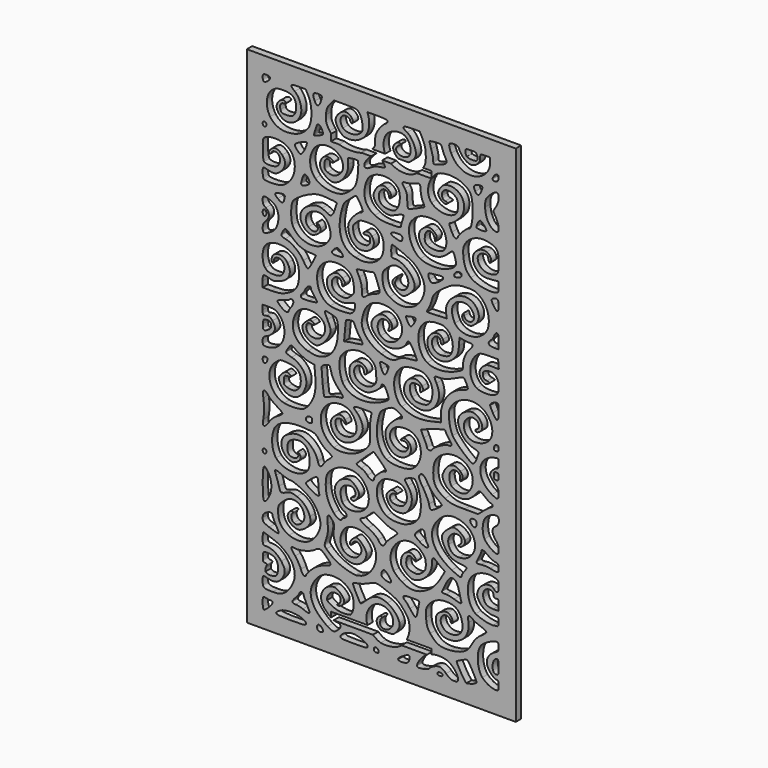
from build123d import *

# Parameters (mm, degrees)
F0_W     = 159.83936
F0_H     = 300
F1_DEPTH = 4


# Not quite as in the source:
# - ends of sketch curves that miss each other by under 0.0002 mm in the source are joined


with BuildPart() as f1:
    # F0 (on Front) → F1 (new body)
    with BuildSketch(Plane.XZ):
        Rectangle(F0_W, F0_H)
        with BuildLine():
            add(Edge.make_bspline(
                [(-66.851123, -137.742915), (-64.379133, -135.200586), (-64.049525, -133.795781), (-65.921818, -133.782129)],
                knots=[0, 0, 0, 0, 1, 1, 1, 1], degree=3))
            add(Edge.make_bspline(
                [(-69.767613, -139.976342), (-69.357941, -139.976342), (-68.045522, -138.971296), (-66.851123, -137.742915)],
                knots=[0, 0, 0, 0, 1, 1, 1, 1], degree=3))
            add(Edge.make_bspline(
                [(-70.512472, -136.460162), (-70.512472, -138.394054), (-70.177285, -139.976342), (-69.767613, -139.976342)],
                knots=[0, 0, 0, 0, 1, 1, 1, 1], degree=3))
            add(Edge.make_bspline(
                [(-68.859836, -133.358345), (-70.416057, -132.968164), (-70.512472, -133.149113), (-70.512472, -136.460162)],
                knots=[0, 0, 0, 0, 1, 1, 1, 1], degree=3))
            add(Edge.make_bspline(
                [(-65.921818, -133.782129), (-66.628778, -133.776572), (-67.950886, -133.586258), (-68.859836, -133.358345)],
                knots=[0, 0, 0, 0, 1, 1, 1, 1], degree=3))
        make_face(mode=Mode.SUBTRACT)
        with BuildLine():
            add(Edge.make_bspline(
                [(-62.339229, -119.598213), (-61.784791, -118.973161), (-61.331159, -117.126303), (-61.331159, -115.494065)],
                knots=[0, 0, 0, 0, 1, 1, 1, 1], degree=3))
            add(Edge.make_bspline(
                [(-68.795819, -119.659993), (-68.196595, -121.120996), (-63.651427, -121.077472), (-62.339229, -119.598213)],
                knots=[0, 0, 0, 0, 1, 1, 1, 1], degree=3))
            add(Edge.make_bspline(
                [(-68.42126, -116.911181), (-68.869686, -117.831987), (-69.038238, -119.06894), (-68.795819, -119.659993)],
                knots=[0, 0, 0, 0, 1, 1, 1, 1], degree=3))
            add(Edge.make_bspline(
                [(-69.101441, -115.236993), (-67.783248, -115.236993), (-67.702605, -115.435478), (-68.42126, -116.911181)],
                knots=[0, 0, 0, 0, 1, 1, 1, 1], degree=3))
            add(Edge.make_bspline(
                [(-70.371078, -112.31638), (-70.568194, -114.865293), (-70.40661, -115.236993), (-69.101441, -115.236993)],
                knots=[0, 0, 0, 0, 1, 1, 1, 1], degree=3))
            add(Edge.make_bspline(
                [(-67.321282, -109.479917), (-70.134768, -109.39607), (-70.146055, -109.406571), (-70.371078, -112.31638)],
                knots=[0, 0, 0, 0, 1, 1, 1, 1], degree=3))
            add(Edge.make_bspline(
                [(-61.331159, -115.494065), (-61.331159, -111.652334), (-63.377855, -109.597429), (-67.321282, -109.479917)],
                knots=[0, 0, 0, 0, 1, 1, 1, 1], degree=3))
        make_face(mode=Mode.SUBTRACT)
        with BuildLine():
            add(Edge.make_bspline(
                [(-57.950885, -127.412999), (-54.596525, -125.305487), (-51.454434, -119.837105), (-51.432503, -116.068621)],
                knots=[0, 0, 0, 0, 1, 1, 1, 1], degree=3))
            add(Edge.make_bspline(
                [(-64.561429, -128.926813), (-61.42975, -128.968088), (-59.850359, -128.606429), (-57.950885, -127.412999)],
                knots=[0, 0, 0, 0, 1, 1, 1, 1], degree=3))
            add(Edge.make_bspline(
                [(-70.512472, -125.064028), (-70.512472, -128.658605), (-70.214078, -128.85228), (-64.561429, -128.926813)],
                knots=[0, 0, 0, 0, 1, 1, 1, 1], degree=3))
            add(Edge.make_bspline(
                [(-68.859836, -122.427958), (-70.405971, -121.979622), (-70.512472, -122.149484), (-70.512472, -125.064028)],
                knots=[0, 0, 0, 0, 1, 1, 1, 1], degree=3))
            add(Edge.make_bspline(
                [(-58.735287, -119.665814), (-61.207531, -123.408372), (-63.40833, -124.008791), (-68.859836, -122.427958)],
                knots=[0, 0, 0, 0, 1, 1, 1, 1], degree=3))
            add(Edge.make_bspline(
                [(-59.480416, -111.241528), (-56.924648, -114.542467), (-56.738809, -116.643476), (-58.735287, -119.665814)],
                knots=[0, 0, 0, 0, 1, 1, 1, 1], degree=3))
            add(Edge.make_bspline(
                [(-68.272484, -106.303345), (-65.025847, -106.303345), (-61.978745, -108.014792), (-59.480416, -111.241528)],
                knots=[0, 0, 0, 0, 1, 1, 1, 1], degree=3))
            add(Edge.make_bspline(
                [(-70.512472, -102.867326), (-70.512472, -106.239419), (-70.470826, -106.303345), (-68.272484, -106.303345)],
                knots=[0, 0, 0, 0, 1, 1, 1, 1], degree=3))
            add(Edge.make_bspline(
                [(-69.979778, -99.431309), (-70.272763, -99.431309), (-70.512472, -100.977518), (-70.512472, -102.867326)],
                knots=[0, 0, 0, 0, 1, 1, 1, 1], degree=3))
            add(Edge.make_bspline(
                [(-64.320321, -101.313195), (-67.140043, -100.278158), (-69.686799, -99.431309), (-69.979778, -99.431309)],
                knots=[0, 0, 0, 0, 1, 1, 1, 1], degree=3))
            add(Edge.make_bspline(
                [(-51.432503, -116.068621), (-51.396697, -109.919845), (-56.362735, -104.23419), (-64.320321, -101.313195)],
                knots=[0, 0, 0, 0, 1, 1, 1, 1], degree=3))
        make_face(mode=Mode.SUBTRACT)
        with BuildLine():
            add(Edge.make_bspline(
                [(-44.804799, -139.191932), (-44.804799, -136.214258), (-55.790918, -134.79281), (-60.045778, -137.219992)],
                knots=[0, 0, 0, 0, 1, 1, 1, 1], degree=3))
            add(Edge.make_bspline(
                [(-53.618858, -140.31993), (-45.936305, -140.31993), (-44.804799, -140.175123), (-44.804799, -139.191932)],
                knots=[0, 0, 0, 0, 1, 1, 1, 1], degree=3))
            add(Edge.make_bspline(
                [(-60.045778, -137.219992), (-64.451981, -139.733507), (-63.236153, -140.31993), (-53.618858, -140.31993)],
                knots=[0, 0, 0, 0, 1, 1, 1, 1], degree=3))
        make_face(mode=Mode.SUBTRACT)
        with BuildLine():
            add(Edge.make_bspline(
                [(-42.608, -132.588884), (-42.611863, -132.30541), (-43.42768, -130.527277), (-44.421293, -128.637464)],
                knots=[0, 0, 0, 0, 1, 1, 1, 1], degree=3))
            add(Edge.make_bspline(
                [(-46.641065, -132.048684), (-44.114874, -133.13091), (-42.598293, -133.334057), (-42.608, -132.588884)],
                knots=[0, 0, 0, 0, 1, 1, 1, 1], degree=3))
            add(Edge.make_bspline(
                [(-50.864464, -131.073668), (-49.753528, -131.090866), (-47.852997, -131.529466), (-46.641065, -132.048684)],
                knots=[0, 0, 0, 0, 1, 1, 1, 1], degree=3))
            add(Edge.make_bspline(
                [(-50.68084, -127.158073), (-53.414736, -130.071294), (-53.459875, -131.033849), (-50.864464, -131.073668)],
                knots=[0, 0, 0, 0, 1, 1, 1, 1], degree=3))
            add(Edge.make_bspline(
                [(-48.477327, -124.146718), (-48.477327, -124.511552), (-49.468908, -125.866642), (-50.68084, -127.158073)],
                knots=[0, 0, 0, 0, 1, 1, 1, 1], degree=3))
            add(Edge.make_bspline(
                [(-46.250839, -124.34243), (-46.277446, -123.346327), (-48.477327, -123.152969), (-48.477327, -124.146718)],
                knots=[0, 0, 0, 0, 1, 1, 1, 1], degree=3))
            add(Edge.make_bspline(
                [(-44.421293, -128.637464), (-45.414915, -126.747651), (-46.238208, -124.814897), (-46.250839, -124.34243)],
                knots=[0, 0, 0, 0, 1, 1, 1, 1], degree=3))
        make_face(mode=Mode.SUBTRACT)
        with BuildLine():
            add(Edge.make_bspline(
                [(-60.96391, -96.752638), (-60.96391, -96.413254), (-61.786246, -94.789737), (-62.791324, -93.144817)],
                knots=[0, 0, 0, 0, 1, 1, 1, 1], degree=3))
            add(Edge.make_bspline(
                [(-66.648158, -95.739437), (-62.272203, -97.402209), (-60.96391, -97.635404), (-60.96391, -96.752638)],
                knots=[0, 0, 0, 0, 1, 1, 1, 1], degree=3))
            add(Edge.make_bspline(
                [(-70.504308, -92.122903), (-70.496926, -94.074753), (-70.134404, -94.414735), (-66.648158, -95.739437)],
                knots=[0, 0, 0, 0, 1, 1, 1, 1], degree=3))
            add(Edge.make_bspline(
                [(-68.702054, -88.858686), (-69.993374, -89.650303), (-70.510131, -90.586243), (-70.504308, -92.122903)],
                knots=[0, 0, 0, 0, 1, 1, 1, 1], degree=3))
            add(Edge.make_bspline(
                [(-64.627584, -88.951449), (-64.638657, -87.44789), (-66.337605, -87.409208), (-68.702054, -88.858686)],
                knots=[0, 0, 0, 0, 1, 1, 1, 1], degree=3))
            add(Edge.make_bspline(
                [(-62.791324, -93.144817), (-63.796402, -91.4999), (-64.62272, -89.612886), (-64.627584, -88.951449)],
                knots=[0, 0, 0, 0, 1, 1, 1, 1], degree=3))
        make_face(mode=Mode.SUBTRACT)
        with BuildLine():
            add(Edge.make_bspline(
                [(-44.804799, -113.864568), (-44.804799, -113.487695), (-43.587869, -111.919092), (-42.100514, -110.37878)],
                knots=[0, 0, 0, 0, 1, 1, 1, 1], degree=3))
            add(Edge.make_bspline(
                [(-45.788993, -114.549791), (-45.24769, -114.549791), (-44.804799, -114.24144), (-44.804799, -113.864568)],
                knots=[0, 0, 0, 0, 1, 1, 1, 1], degree=3))
            add(Edge.make_bspline(
                [(-47.799657, -111.639848), (-47.2351, -113.240318), (-46.330299, -114.549791), (-45.788993, -114.549791)],
                knots=[0, 0, 0, 0, 1, 1, 1, 1], degree=3))
            add(Edge.make_bspline(
                [(-51.222492, -105.792667), (-49.904492, -107.408147), (-48.36422, -110.039375), (-47.799657, -111.639848)],
                knots=[0, 0, 0, 0, 1, 1, 1, 1], degree=3))
            add(Edge.make_bspline(
                [(-51.427574, -101.834003), (-54.273319, -101.249226), (-54.228841, -102.107776), (-51.222492, -105.792667)],
                knots=[0, 0, 0, 0, 1, 1, 1, 1], degree=3))
            add(Edge.make_bspline(
                [(-39.479533, -98.756388), (-42.077503, -100.668347), (-48.743852, -102.385495), (-51.427574, -101.834003)],
                knots=[0, 0, 0, 0, 1, 1, 1, 1], degree=3))
            add(Edge.make_bspline(
                [(-32.834535, -99.975684), (-35.946379, -96.994099), (-36.857713, -96.826875), (-39.479533, -98.756388)],
                knots=[0, 0, 0, 0, 1, 1, 1, 1], degree=3))
            add(Edge.make_bspline(
                [(-32.134591, -104.66976), (-29.441323, -104.064126), (-29.586973, -103.087313), (-32.834535, -99.975684)],
                knots=[0, 0, 0, 0, 1, 1, 1, 1], degree=3))
            add(Edge.make_bspline(
                [(-42.100514, -110.37878), (-39.353689, -107.534184), (-35.787246, -105.491127), (-32.134591, -104.66976)],
                knots=[0, 0, 0, 0, 1, 1, 1, 1], degree=3))
        make_face(mode=Mode.SUBTRACT)
        with BuildLine():
            add(Edge.make_bspline(
                [(-42.534711, -95.263732), (-39.457316, -93.21355), (-36.778772, -88.993237), (-36.245753, -85.354854)],
                knots=[0, 0, 0, 0, 1, 1, 1, 1], degree=3))
            add(Edge.make_bspline(
                [(-54.793282, -96.101009), (-51.039853, -97.746627), (-45.715809, -97.382984), (-42.534711, -95.263732)],
                knots=[0, 0, 0, 0, 1, 1, 1, 1], degree=3))
            add(Edge.make_bspline(
                [(-61.331159, -86.153305), (-61.331159, -91.034749), (-59.30013, -94.125056), (-54.793282, -96.101009)],
                knots=[0, 0, 0, 0, 1, 1, 1, 1], degree=3))
            add(Edge.make_bspline(
                [(-58.237959, -79.453068), (-61.187942, -82.027573), (-61.331159, -82.337805), (-61.331159, -86.153305)],
                knots=[0, 0, 0, 0, 1, 1, 1, 1], degree=3))
            add(Edge.make_bspline(
                [(-52.512159, -76.753564), (-54.560883, -76.753564), (-55.830779, -77.352277), (-58.237959, -79.453068)],
                knots=[0, 0, 0, 0, 1, 1, 1, 1], degree=3))
            add(Edge.make_bspline(
                [(-48.713504, -88.43603), (-43.126597, -85.489736), (-45.967235, -76.753564), (-52.512159, -76.753564)],
                knots=[0, 0, 0, 0, 1, 1, 1, 1], degree=3))
            add(Edge.make_bspline(
                [(-51.959886, -88.70945), (-50.982304, -89.282646), (-50.1928, -89.216154), (-48.713504, -88.43603)],
                knots=[0, 0, 0, 0, 1, 1, 1, 1], degree=3))
            add(Edge.make_bspline(
                [(-52.850801, -83.931385), (-54.027847, -85.258299), (-53.559198, -87.771711), (-51.959886, -88.70945)],
                knots=[0, 0, 0, 0, 1, 1, 1, 1], degree=3))
            add(Edge.make_bspline(
                [(-53.177417, -82.938404), (-52.20786, -82.938404), (-52.143511, -83.134034), (-52.850801, -83.931385)],
                knots=[0, 0, 0, 0, 1, 1, 1, 1], degree=3))
            add(Edge.make_bspline(
                [(-55.252671, -84.720356), (-54.775373, -83.740297), (-53.841512, -82.938404), (-53.177417, -82.938404)],
                knots=[0, 0, 0, 0, 1, 1, 1, 1], degree=3))
            add(Edge.make_bspline(
                [(-51.698981, -90.927193), (-54.873484, -89.716311), (-56.393111, -87.062152), (-55.252671, -84.720356)],
                knots=[0, 0, 0, 0, 1, 1, 1, 1], degree=3))
            add(Edge.make_bspline(
                [(-46.924696, -90.555485), (-49.065924, -91.626569), (-49.729941, -91.678263), (-51.698981, -90.927193)],
                knots=[0, 0, 0, 0, 1, 1, 1, 1], degree=3))
            add(Edge.make_bspline(
                [(-43.0524, -87.104162), (-43.81423, -88.318121), (-45.556766, -89.871214), (-46.924696, -90.555485)],
                knots=[0, 0, 0, 0, 1, 1, 1, 1], degree=3))
            add(Edge.make_bspline(
                [(-42.521087, -82.230622), (-41.785202, -84.528618), (-41.858595, -85.201866), (-43.0524, -87.104162)],
                knots=[0, 0, 0, 0, 1, 1, 1, 1], degree=3))
            add(Edge.make_bspline(
                [(-50.222023, -74.344509), (-46.485414, -75.679639), (-43.708159, -78.523664), (-42.521087, -82.230622)],
                knots=[0, 0, 0, 0, 1, 1, 1, 1], degree=3))
            add(Edge.make_bspline(
                [(-56.166876, -74.295186), (-53.627402, -73.302458), (-53.126918, -73.306618), (-50.222023, -74.344509)],
                knots=[0, 0, 0, 0, 1, 1, 1, 1], degree=3))
            add(Edge.make_bspline(
                [(-59.525114, -75.379176), (-59.203192, -75.379176), (-57.691983, -74.891382), (-56.166876, -74.295186)],
                knots=[0, 0, 0, 0, 1, 1, 1, 1], degree=3))
            add(Edge.make_bspline(
                [(-60.834845, -72.458557), (-60.436422, -74.064898), (-59.847043, -75.379176), (-59.525114, -75.379176)],
                knots=[0, 0, 0, 0, 1, 1, 1, 1], degree=3))
            add(Edge.make_bspline(
                [(-62.513791, -67.33076), (-61.988798, -68.544708), (-61.233274, -70.852218), (-60.834845, -72.458557)],
                knots=[0, 0, 0, 0, 1, 1, 1, 1], degree=3))
            add(Edge.make_bspline(
                [(-62.988957, -64.675073), (-63.252608, -64.921744), (-63.038812, -66.116809), (-62.513791, -67.33076)],
                knots=[0, 0, 0, 0, 1, 1, 1, 1], degree=3))
            add(Edge.make_bspline(
                [(-59.301337, -65.679656), (-61.065878, -64.880467), (-62.725307, -64.428402), (-62.988957, -64.675073)],
                knots=[0, 0, 0, 0, 1, 1, 1, 1], degree=3))
            add(Edge.make_bspline(
                [(-54.097048, -67.13273), (-55.194861, -67.13273), (-57.536795, -66.478849), (-59.301337, -65.679656)],
                knots=[0, 0, 0, 0, 1, 1, 1, 1], degree=3))
            add(Edge.make_bspline(
                [(-42.29059, -72.676084), (-45.647849, -69.918199), (-51.580458, -67.13273), (-54.097048, -67.13273)],
                knots=[0, 0, 0, 0, 1, 1, 1, 1], degree=3))
            add(Edge.make_bspline(
                [(-36.245753, -85.354854), (-35.688252, -81.549402), (-38.391817, -75.878807), (-42.29059, -72.676084)],
                knots=[0, 0, 0, 0, 1, 1, 1, 1], degree=3))
        make_face(mode=Mode.SUBTRACT)
        with BuildLine():
            add(Edge.make_bspline(
                [(-34.521736, -139.770179), (-34.521736, -138.620961), (-36.011083, -137.227506), (-37.239401, -137.227506)],
                knots=[0, 0, 0, 0, 1, 1, 1, 1], degree=3))
            add(Edge.make_bspline(
                [(-37.704586, -140.205392), (-36.842057, -141.012397), (-34.521736, -140.695109), (-34.521736, -139.770179)],
                knots=[0, 0, 0, 0, 1, 1, 1, 1], degree=3))
            add(Edge.make_bspline(
                [(-37.239401, -137.227506), (-38.227995, -137.227506), (-38.567117, -139.398413), (-37.704586, -140.205392)],
                knots=[0, 0, 0, 0, 1, 1, 1, 1], degree=3))
        make_face(mode=Mode.SUBTRACT)
        with BuildLine():
            add(Edge.make_bspline(
                [(-8.07955, -139.178623), (-8.07955, -137.396337), (-14.207168, -134.924335), (-17.576935, -135.347218)],
                knots=[0, 0, 0, 0, 1, 1, 1, 1], degree=3))
            add(Edge.make_bspline(
                [(-16.159107, -140.31993), (-9.119291, -140.31993), (-8.07955, -140.17306), (-8.07955, -139.178623)],
                knots=[0, 0, 0, 0, 1, 1, 1, 1], degree=3))
            add(Edge.make_bspline(
                [(-24.238662, -139.19635), (-24.238662, -140.168218), (-23.14774, -140.31993), (-16.159107, -140.31993)],
                knots=[0, 0, 0, 0, 1, 1, 1, 1], degree=3))
            add(Edge.make_bspline(
                [(-17.576935, -135.347218), (-20.959281, -135.771663), (-24.238662, -137.666476), (-24.238662, -139.19635)],
                knots=[0, 0, 0, 0, 1, 1, 1, 1], degree=3))
        make_face(mode=Mode.SUBTRACT)
        with BuildLine():
            add(Edge.make_bspline(
                [(-1.607212, -139.468818), (-1.975941, -137.677457), (-4.40703, -137.47767), (-4.40703, -139.238736)],
                knots=[0, 0, 0, 0, 1, 1, 1, 1], degree=3))
            add(Edge.make_bspline(
                [(-2.88416, -140.663544), (-1.833015, -140.663544), (-1.437468, -140.293471), (-1.607212, -139.468818)],
                knots=[0, 0, 0, 0, 1, 1, 1, 1], degree=3))
            add(Edge.make_bspline(
                [(-4.40703, -139.238736), (-4.40703, -140.222193), (-3.935312, -140.663544), (-2.88416, -140.663544)],
                knots=[0, 0, 0, 0, 1, 1, 1, 1], degree=3))
        make_face(mode=Mode.SUBTRACT)
        with BuildLine():
            add(Edge.make_bspline(
                [(-12.375275, -103.537076), (-6.816897, -102.092623), (-2.310755, -94.8983), (-3.177506, -88.852301)],
                knots=[0, 0, 0, 0, 1, 1, 1, 1], degree=3))
            add(Edge.make_bspline(
                [(-15.424603, -104.180302), (-15.222612, -104.209835), (-13.850411, -103.920425), (-12.375275, -103.537076)],
                knots=[0, 0, 0, 0, 1, 1, 1, 1], degree=3))
            add(Edge.make_bspline(
                [(-32.618966, -96.064044), (-28.45692, -100.366878), (-22.604916, -103.129205), (-15.424603, -104.180302)],
                knots=[0, 0, 0, 0, 1, 1, 1, 1], degree=3))
            add(Edge.make_bspline(
                [(-32.69614, -90.777262), (-33.95249, -94.514295), (-33.94995, -94.688036), (-32.618966, -96.064044)],
                knots=[0, 0, 0, 0, 1, 1, 1, 1], degree=3))
            add(Edge.make_bspline(
                [(-31.878117, -82.520619), (-31.517672, -85.812202), (-31.722714, -87.881791), (-32.69614, -90.777262)],
                knots=[0, 0, 0, 0, 1, 1, 1, 1], degree=3))
            add(Edge.make_bspline(
                [(-29.132991, -79.903929), (-31.547867, -76.802023), (-32.41393, -77.627568), (-31.878117, -82.520619)],
                knots=[0, 0, 0, 0, 1, 1, 1, 1], degree=3))
            add(Edge.make_bspline(
                [(-28.275585, -84.980614), (-27.884044, -82.317085), (-28.058507, -81.284104), (-29.132991, -79.903929)],
                knots=[0, 0, 0, 0, 1, 1, 1, 1], degree=3))
            add(Edge.make_bspline(
                [(-13.347211, -97.774321), (-20.387766, -101.180668), (-29.508038, -93.364535), (-28.275585, -84.980614)],
                knots=[0, 0, 0, 0, 1, 1, 1, 1], degree=3))
            add(Edge.make_bspline(
                [(-8.81406, -90.806667), (-8.81406, -93.535064), (-10.756689, -96.520979), (-13.347211, -97.774321)],
                knots=[0, 0, 0, 0, 1, 1, 1, 1], degree=3))
            add(Edge.make_bspline(
                [(-14.650035, -84.312824), (-12.98112, -84.312824), (-8.81406, -88.949623), (-8.81406, -90.806667)],
                knots=[0, 0, 0, 0, 1, 1, 1, 1], degree=3))
            add(Edge.make_bspline(
                [(-18.627659, -88.781052), (-19.107537, -87.611062), (-16.17144, -84.312824), (-14.650035, -84.312824)],
                knots=[0, 0, 0, 0, 1, 1, 1, 1], degree=3))
            add(Edge.make_bspline(
                [(-17.331227, -88.309895), (-18.033223, -89.627284), (-18.248495, -89.705519), (-18.627659, -88.781052)],
                knots=[0, 0, 0, 0, 1, 1, 1, 1], degree=3))
            add(Edge.make_bspline(
                [(-12.942988, -87.420001), (-14.493277, -85.96955), (-16.276863, -86.331243), (-17.331227, -88.309895)],
                knots=[0, 0, 0, 0, 1, 1, 1, 1], degree=3))
            add(Edge.make_bspline(
                [(-13.274398, -93.4974), (-11.447971, -91.325002), (-11.317936, -88.940397), (-12.942988, -87.420001)],
                knots=[0, 0, 0, 0, 1, 1, 1, 1], degree=3))
            add(Edge.make_bspline(
                [(-22.435786, -93.621307), (-19.85114, -96.039509), (-15.360598, -95.978774), (-13.274398, -93.4974)],
                knots=[0, 0, 0, 0, 1, 1, 1, 1], degree=3))
            add(Edge.make_bspline(
                [(-19.92597, -80.578847), (-24.285623, -82.688124), (-25.786305, -90.486561), (-22.435786, -93.621307)],
                knots=[0, 0, 0, 0, 1, 1, 1, 1], degree=3))
            add(Edge.make_bspline(
                [(-3.177506, -88.852301), (-4.20483, -81.686316), (-13.116296, -77.284197), (-19.92597, -80.578847)],
                knots=[0, 0, 0, 0, 1, 1, 1, 1], degree=3))
        make_face(mode=Mode.SUBTRACT)
        with BuildLine():
            add(Edge.make_bspline(
                [(2.532647, -81.632981), (3.138394, -80.537029), (4.964781, -78.574602), (6.591284, -77.272034)],
                knots=[0, 0, 0, 0, 1, 1, 1, 1], degree=3))
            add(Edge.make_bspline(
                [(-1.845845, -81.365733), (-0.002744, -84.116739), (1.121896, -84.185385), (2.532647, -81.632981)],
                knots=[0, 0, 0, 0, 1, 1, 1, 1], degree=3))
            add(Edge.make_bspline(
                [(-7.886904, -77.097184), (-4.96047, -78.419537), (-2.794244, -79.95017), (-1.845845, -81.365733)],
                knots=[0, 0, 0, 0, 1, 1, 1, 1], degree=3))
            add(Edge.make_bspline(
                [(-11.062806, -72.987398), (-13.548752, -73.725588), (-12.58316, -74.975109), (-7.886904, -77.097184)],
                knots=[0, 0, 0, 0, 1, 1, 1, 1], degree=3))
            add(Edge.make_bspline(
                [(-7.412723, -70.192271), (-8.637194, -71.497058), (-10.279732, -72.754858), (-11.062806, -72.987398)],
                knots=[0, 0, 0, 0, 1, 1, 1, 1], degree=3))
            add(Edge.make_bspline(
                [(-4.411761, -67.819932), (-4.837822, -67.819932), (-6.188253, -68.887481), (-7.412723, -70.192271)],
                knots=[0, 0, 0, 0, 1, 1, 1, 1], degree=3))
            add(Edge.make_bspline(
                [(0.108648, -70.23063), (-1.951522, -68.904747), (-3.985702, -67.819932), (-4.411761, -67.819932)],
                knots=[0, 0, 0, 0, 1, 1, 1, 1], degree=3))
            add(Edge.make_bspline(
                [(6.701483, -73.067276), (5.135594, -72.833003), (2.168821, -71.556515), (0.108648, -70.23063)],
                knots=[0, 0, 0, 0, 1, 1, 1, 1], degree=3))
            add(Edge.make_bspline(
                [(9.548566, -74.198475), (9.548566, -73.810588), (8.267382, -73.301546), (6.701483, -73.067276)],
                knots=[0, 0, 0, 0, 1, 1, 1, 1], degree=3))
            add(Edge.make_bspline(
                [(6.591284, -77.272034), (8.217786, -75.969466), (9.548566, -74.586368), (9.548566, -74.198475)],
                knots=[0, 0, 0, 0, 1, 1, 1, 1], degree=3))
        make_face(mode=Mode.SUBTRACT)
        with BuildLine():
            add(Edge.make_bspline(
                [(-66.975198, -80.26784), (-64.811809, -76.666487), (-64.811809, -71.343047), (-66.975198, -67.741695)],
                knots=[0, 0, 0, 0, 1, 1, 1, 1], degree=3))
            add(Edge.make_bspline(
                [(-70.512472, -74.004766), (-70.512472, -83.916674), (-69.860535, -85.07099), (-66.975198, -80.26784)],
                knots=[0, 0, 0, 0, 1, 1, 1, 1], degree=3))
            add(Edge.make_bspline(
                [(-66.975198, -67.741695), (-69.860535, -62.938547), (-70.512472, -64.092863), (-70.512472, -74.004766)],
                knots=[0, 0, 0, 0, 1, 1, 1, 1], degree=3))
        make_face(mode=Mode.SUBTRACT)
        with BuildLine():
            add(Edge.make_bspline(
                [(-68.308958, -56.824674), (-68.308958, -56.061116), (-68.798628, -55.450264), (-69.410715, -55.450264)],
                knots=[0, 0, 0, 0, 1, 1, 1, 1], degree=3))
            add(Edge.make_bspline(
                [(-69.410715, -58.199079), (-68.798628, -58.199079), (-68.308958, -57.588233), (-68.308958, -56.824674)],
                knots=[0, 0, 0, 0, 1, 1, 1, 1], degree=3))
            add(Edge.make_bspline(
                [(-70.512472, -56.824674), (-70.512472, -57.588233), (-70.022802, -58.199079), (-69.410715, -58.199079)],
                knots=[0, 0, 0, 0, 1, 1, 1, 1], degree=3))
            add(Edge.make_bspline(
                [(-69.410715, -55.450264), (-70.022802, -55.450264), (-70.512472, -56.061116), (-70.512472, -56.824674)],
                knots=[0, 0, 0, 0, 1, 1, 1, 1], degree=3))
        make_face(mode=Mode.SUBTRACT)
        with BuildLine():
            add(Edge.make_bspline(
                [(-36.996804, -68.335335), (-37.240393, -67.484922), (-37.444207, -65.320228), (-37.449721, -63.524911)],
                knots=[0, 0, 0, 0, 1, 1, 1, 1], degree=3))
            add(Edge.make_bspline(
                [(-37.924963, -69.840235), (-36.855041, -69.872448), (-36.65119, -69.541949), (-36.996804, -68.335335)],
                knots=[0, 0, 0, 0, 1, 1, 1, 1], degree=3))
            add(Edge.make_bspline(
                [(-44.804799, -65.674595), (-44.804799, -66.567977), (-39.477715, -69.793451), (-37.924963, -69.840235)],
                knots=[0, 0, 0, 0, 1, 1, 1, 1], degree=3))
            add(Edge.make_bspline(
                [(-38.377884, -60.279286), (-39.440642, -60.30077), (-44.804799, -64.803944), (-44.804799, -65.674595)],
                knots=[0, 0, 0, 0, 1, 1, 1, 1], degree=3))
            add(Edge.make_bspline(
                [(-37.449721, -63.524911), (-37.456335, -61.36662), (-37.770816, -60.266993), (-38.377884, -60.279286)],
                knots=[0, 0, 0, 0, 1, 1, 1, 1], degree=3))
        make_face(mode=Mode.SUBTRACT)
        with BuildLine():
            add(Edge.make_bspline(
                [(-47.01643, -61.295423), (-43.782782, -59.730926), (-42.601285, -57.656966), (-42.601285, -53.545217)],
                knots=[0, 0, 0, 0, 1, 1, 1, 1], degree=3))
            add(Edge.make_bspline(
                [(-62.55736, -58.199071), (-59.61986, -61.99177), (-51.712141, -63.567289), (-47.01643, -61.295423)],
                knots=[0, 0, 0, 0, 1, 1, 1, 1], degree=3))
            add(Edge.make_bspline(
                [(-62.205095, -41.108231), (-65.633753, -44.581374), (-65.827414, -53.977009), (-62.55736, -58.199071)],
                knots=[0, 0, 0, 0, 1, 1, 1, 1], degree=3))
            add(Edge.make_bspline(
                [(-42.395135, -37.32525), (-51.658557, -36.137319), (-58.60794, -37.4644), (-62.205095, -41.108231)],
                knots=[0, 0, 0, 0, 1, 1, 1, 1], degree=3))
            add(Edge.make_bspline(
                [(-36.844857, -40.622308), (-38.72283, -38.175677), (-39.537561, -37.691701), (-42.395135, -37.32525)],
                knots=[0, 0, 0, 0, 1, 1, 1, 1], degree=3))
            add(Edge.make_bspline(
                [(-32.011991, -44.815909), (-33.459476, -44.086587), (-35.634266, -42.199471), (-36.844857, -40.622308)],
                knots=[0, 0, 0, 0, 1, 1, 1, 1], degree=3))
            add(Edge.make_bspline(
                [(-29.380196, -46.717247), (-29.380196, -46.400834), (-30.564503, -45.54523), (-32.011991, -44.815909)],
                knots=[0, 0, 0, 0, 1, 1, 1, 1], degree=3))
            add(Edge.make_bspline(
                [(-31.421483, -48.899565), (-30.298777, -48.0157), (-29.380196, -47.033662), (-29.380196, -46.717247)],
                knots=[0, 0, 0, 0, 1, 1, 1, 1], degree=3))
            add(Edge.make_bspline(
                [(-34.48362, -52.291213), (-33.922153, -51.309659), (-32.54419, -49.783418), (-31.421483, -48.899565)],
                knots=[0, 0, 0, 0, 1, 1, 1, 1], degree=3))
            add(Edge.make_bspline(
                [(-37.75115, -51.853677), (-37.177763, -54.535978), (-35.867999, -54.71136), (-34.48362, -52.291213)],
                knots=[0, 0, 0, 0, 1, 1, 1, 1], degree=3))
            add(Edge.make_bspline(
                [(-49.460121, -41.706179), (-44.704082, -41.706179), (-38.832597, -46.794664), (-37.75115, -51.853677)],
                knots=[0, 0, 0, 0, 1, 1, 1, 1], degree=3))
            add(Edge.make_bspline(
                [(-57.95803, -45.561176), (-56.261539, -43.543324), (-52.211754, -41.706179), (-49.460121, -41.706179)],
                knots=[0, 0, 0, 0, 1, 1, 1, 1], degree=3))
            add(Edge.make_bspline(
                [(-55.075436, -56.487076), (-59.321626, -54.432693), (-60.777455, -48.914664), (-57.95803, -45.561176)],
                knots=[0, 0, 0, 0, 1, 1, 1, 1], degree=3))
            add(Edge.make_bspline(
                [(-50.732892, -56.506259), (-52.658726, -57.438007), (-53.114138, -57.435994), (-55.075436, -56.487076)],
                knots=[0, 0, 0, 0, 1, 1, 1, 1], degree=3))
            add(Edge.make_bspline(
                [(-48.872553, -51.422211), (-47.155976, -52.931394), (-47.97601, -55.172423), (-50.732892, -56.506259)],
                knots=[0, 0, 0, 0, 1, 1, 1, 1], degree=3))
            add(Edge.make_bspline(
                [(-49.635141, -51.161392), (-49.92011, -50.685555), (-49.576945, -50.802924), (-48.872553, -51.422211)],
                knots=[0, 0, 0, 0, 1, 1, 1, 1], degree=3))
            add(Edge.make_bspline(
                [(-52.052446, -54.763062), (-49.939059, -54.763062), (-48.638579, -52.825404), (-49.635141, -51.161392)],
                knots=[0, 0, 0, 0, 1, 1, 1, 1], degree=3))
            add(Edge.make_bspline(
                [(-55.822373, -50.800821), (-55.822373, -53.604153), (-54.719718, -54.763062), (-52.052446, -54.763062)],
                knots=[0, 0, 0, 0, 1, 1, 1, 1], degree=3))
            add(Edge.make_bspline(
                [(-51.745039, -45.130607), (-54.7624, -46.0623), (-55.822373, -47.536373), (-55.822373, -50.800821)],
                knots=[0, 0, 0, 0, 1, 1, 1, 1], degree=3))
            add(Edge.make_bspline(
                [(-42.601285, -53.545217), (-42.601285, -46.848769), (-46.29649, -43.44823), (-51.745039, -45.130607)],
                knots=[0, 0, 0, 0, 1, 1, 1, 1], degree=3))
        make_face(mode=Mode.SUBTRACT)
        with BuildLine():
            add(Edge.make_bspline(
                [(-66.721645, -40.709353), (-65.61434, -39.001293), (-63.467643, -36.999961), (-61.769394, -36.092445)],
                knots=[0, 0, 0, 0, 1, 1, 1, 1], degree=3))
            add(Edge.make_bspline(
                [(-70.164427, -40.503584), (-70.871519, -44.784931), (-69.420014, -44.871683), (-66.721645, -40.709353)],
                knots=[0, 0, 0, 0, 1, 1, 1, 1], degree=3))
            add(Edge.make_bspline(
                [(-70.121514, -29.16472), (-69.424057, -33.810509), (-69.432612, -36.072588), (-70.164427, -40.503584)],
                knots=[0, 0, 0, 0, 1, 1, 1, 1], degree=3))
            add(Edge.make_bspline(
                [(-66.979671, -27.245072), (-69.675902, -23.833069), (-70.817246, -24.530424), (-70.121514, -29.16472)],
                knots=[0, 0, 0, 0, 1, 1, 1, 1], degree=3))
            add(Edge.make_bspline(
                [(-62.06726, -31.089987), (-63.886035, -30.092754), (-66.096618, -28.362537), (-66.979671, -27.245072)],
                knots=[0, 0, 0, 0, 1, 1, 1, 1], degree=3))
            add(Edge.make_bspline(
                [(-58.766053, -33.696844), (-58.762749, -33.260303), (-60.248485, -32.08722), (-62.06726, -31.089987)],
                knots=[0, 0, 0, 0, 1, 1, 1, 1], degree=3))
            add(Edge.make_bspline(
                [(-61.769394, -36.092445), (-60.120664, -35.211407), (-58.76916, -34.133378), (-58.766053, -33.696844)],
                knots=[0, 0, 0, 0, 1, 1, 1, 1], degree=3))
        make_face(mode=Mode.SUBTRACT)
        with BuildLine():
            add(Edge.make_bspline(
                [(-68.020292, -9.695006), (-67.27535, -7.878737), (-67.507402, -7.345995), (-69.043461, -7.345995)],
                knots=[0, 0, 0, 0, 1, 1, 1, 1], degree=3))
            add(Edge.make_bspline(
                [(-70.512472, -9.064009), (-70.512472, -10.982503), (-68.733134, -11.433017), (-68.020292, -9.695006)],
                knots=[0, 0, 0, 0, 1, 1, 1, 1], degree=3))
            add(Edge.make_bspline(
                [(-69.043461, -7.345995), (-70.120737, -7.345995), (-70.512472, -7.804137), (-70.512472, -9.064009)],
                knots=[0, 0, 0, 0, 1, 1, 1, 1], degree=3))
        make_face(mode=Mode.SUBTRACT)
        with BuildLine():
            add(Edge.make_bspline(
                [(-41.132279, -31.741735), (-41.132279, -29.974757), (-41.628555, -29.717625), (-43.642968, -30.440847)],
                knots=[0, 0, 0, 0, 1, 1, 1, 1], degree=3))
            add(Edge.make_bspline(
                [(-42.96854, -33.459743), (-41.499528, -33.459743), (-41.132279, -33.116139), (-41.132279, -31.741735)],
                knots=[0, 0, 0, 0, 1, 1, 1, 1], degree=3))
            add(Edge.make_bspline(
                [(-43.642968, -30.440847), (-45.598858, -31.143054), (-45.081302, -33.459743), (-42.96854, -33.459743)],
                knots=[0, 0, 0, 0, 1, 1, 1, 1], degree=3))
        make_face(mode=Mode.SUBTRACT)
        with BuildLine():
            Line((-39.781068, -2.006402), (-39.278005, -7.65669))
            add(Edge.make_bspline(
                [(-39.627284, -17.148279), (-39.098064, -14.763211), (-38.965651, -11.164962), (-39.278005, -7.65669)],
                knots=[0, 0, 0, 0, 1, 1, 1, 1], degree=3))
            add(Edge.make_bspline(
                [(-46.271789, -27.273899), (-43.678396, -25.975337), (-40.516877, -21.157468), (-39.627284, -17.148279)],
                knots=[0, 0, 0, 0, 1, 1, 1, 1], degree=3))
            add(Edge.make_bspline(
                [(-57.786608, -27.895995), (-54.240503, -28.684078), (-48.464936, -28.372041), (-46.271789, -27.273899)],
                knots=[0, 0, 0, 0, 1, 1, 1, 1], degree=3))
            add(Edge.make_bspline(
                [(-62.788167, -8.147011), (-69.589921, -13.978938), (-66.559075, -25.946426), (-57.786608, -27.895995)],
                knots=[0, 0, 0, 0, 1, 1, 1, 1], degree=3))
            add(Edge.make_bspline(
                [(-56.078047, -6.123491), (-59.799078, -5.834783), (-60.250021, -5.970773), (-62.788167, -8.147011)],
                knots=[0, 0, 0, 0, 1, 1, 1, 1], degree=3))
            add(Edge.make_bspline(
                [(-47.883604, -12.45683), (-48.173807, -8.286338), (-50.402475, -6.563842), (-56.078047, -6.123491)],
                knots=[0, 0, 0, 0, 1, 1, 1, 1], degree=3))
            add(Edge.make_bspline(
                [(-56.106439, -19.058052), (-51.143297, -20.823524), (-47.504673, -17.902458), (-47.883604, -12.45683)],
                knots=[0, 0, 0, 0, 1, 1, 1, 1], degree=3))
            add(Edge.make_bspline(
                [(-57.88668, -15.765452), (-58.087068, -18.031029), (-57.8712, -18.430307), (-56.106439, -19.058052)],
                knots=[0, 0, 0, 0, 1, 1, 1, 1], degree=3))
            add(Edge.make_bspline(
                [(-55.638749, -13.214321), (-57.449013, -13.190059), (-57.682304, -13.454799), (-57.88668, -15.765452)],
                knots=[0, 0, 0, 0, 1, 1, 1, 1], degree=3))
            add(Edge.make_bspline(
                [(-55.107839, -11.459221), (-53.02744, -12.50092), (-53.252921, -13.246317), (-55.638749, -13.214321)],
                knots=[0, 0, 0, 0, 1, 1, 1, 1], degree=3))
            add(Edge.make_bspline(
                [(-58.780365, -12.756587), (-56.952737, -11.046662), (-56.354114, -10.835185), (-55.107839, -11.459221)],
                knots=[0, 0, 0, 0, 1, 1, 1, 1], degree=3))
            add(Edge.make_bspline(
                [(-60.96391, -15.91731), (-60.96391, -15.302527), (-59.981314, -13.880201), (-58.780365, -12.756587)],
                knots=[0, 0, 0, 0, 1, 1, 1, 1], degree=3))
            add(Edge.make_bspline(
                [(-56.455217, -22.170065), (-58.750799, -21.059424), (-60.96391, -17.99023), (-60.96391, -15.91731)],
                knots=[0, 0, 0, 0, 1, 1, 1, 1], degree=3))
            add(Edge.make_bspline(
                [(-44.851426, -15.102168), (-46.684772, -21.549998), (-51.577336, -24.530074), (-56.455217, -22.170065)],
                knots=[0, 0, 0, 0, 1, 1, 1, 1], degree=3))
            add(Edge.make_bspline(
                [(-53.314421, -2.51912), (-47.26899, -4.10273), (-43.371567, -9.897539), (-44.851426, -15.102168)],
                knots=[0, 0, 0, 0, 1, 1, 1, 1], degree=3))
            add(Edge.make_bspline(
                [(-56.556881, -1.006084), (-56.556881, -1.371095), (-55.097775, -2.051963), (-53.314421, -2.51912)],
                knots=[0, 0, 0, 0, 1, 1, 1, 1], degree=3))
            add(Edge.make_bspline(
                [(-53.534304, 3.649262), (-54.14097, 3.649262), (-56.556881, -0.071705), (-56.556881, -1.006084)],
                knots=[0, 0, 0, 0, 1, 1, 1, 1], degree=3))
            add(Edge.make_bspline(
                [(-49.205746, 1.240218), (-51.31017, 2.565196), (-53.258022, 3.649262), (-53.534304, 3.649262)],
                knots=[0, 0, 0, 0, 1, 1, 1, 1], degree=3))
            add(Edge.make_bspline(
                [(-42.580291, -1.587617), (-44.119864, -1.357284), (-47.101319, -0.084754), (-49.205746, 1.240218)],
                knots=[0, 0, 0, 0, 1, 1, 1, 1], degree=3))
            Line((-42.580291, -1.587617), (-39.781068, -2.006402))
        make_face(mode=Mode.SUBTRACT)
        with BuildLine():
            add(Edge.make_bspline(
                [(-23.504158, -77.487095), (-23.504158, -77.134601), (-22.843104, -76.649901), (-22.035146, -76.409982)],
                knots=[0, 0, 0, 0, 1, 1, 1, 1], degree=3))
            add(Edge.make_bspline(
                [(-28.204089, -75.875034), (-26.510893, -77.951984), (-23.504144, -78.983285), (-23.504158, -77.487095)],
                knots=[0, 0, 0, 0, 1, 1, 1, 1], degree=3))
            add(Edge.make_bspline(
                [(-33.036569, -62.771933), (-33.019265, -67.815273), (-31.569089, -71.747399), (-28.204089, -75.875034)],
                knots=[0, 0, 0, 0, 1, 1, 1, 1], degree=3))
            add(Edge.make_bspline(
                [(-27.719692, -52.392364), (-32.059409, -55.303106), (-33.055513, -57.247685), (-33.036569, -62.771933)],
                knots=[0, 0, 0, 0, 1, 1, 1, 1], degree=3))
            add(Edge.make_bspline(
                [(-14.111306, -50.908096), (-17.678173, -49.182372), (-23.954428, -49.866931), (-27.719692, -52.392364)],
                knots=[0, 0, 0, 0, 1, 1, 1, 1], degree=3))
            add(Edge.make_bspline(
                [(-8.585349, -66.433195), (-5.737905, -61.311883), (-8.469416, -53.637741), (-14.111306, -50.908096)],
                knots=[0, 0, 0, 0, 1, 1, 1, 1], degree=3))
            add(Edge.make_bspline(
                [(-23.135056, -68.510444), (-20.768493, -72.792146), (-11.375295, -71.451089), (-8.585349, -66.433195)],
                knots=[0, 0, 0, 0, 1, 1, 1, 1], degree=3))
            add(Edge.make_bspline(
                [(-23.532206, -60.996968), (-24.572966, -62.816407), (-24.392216, -66.235919), (-23.135056, -68.510444)],
                knots=[0, 0, 0, 0, 1, 1, 1, 1], degree=3))
            add(Edge.make_bspline(
                [(-16.960229, -58.852912), (-18.828049, -57.917663), (-22.445941, -59.097971), (-23.532206, -60.996968)],
                knots=[0, 0, 0, 0, 1, 1, 1, 1], degree=3))
            add(Edge.make_bspline(
                [(-16.967505, -63.913907), (-14.839284, -63.393204), (-14.834299, -59.91741), (-16.960229, -58.852912)],
                knots=[0, 0, 0, 0, 1, 1, 1, 1], degree=3))
            add(Edge.make_bspline(
                [(-16.850249, -65.758322), (-18.33158, -65.758322), (-18.426142, -64.270787), (-16.967505, -63.913907)],
                knots=[0, 0, 0, 0, 1, 1, 1, 1], degree=3))
            add(Edge.make_bspline(
                [(-13.221079, -61.238636), (-13.221079, -62.964013), (-15.464822, -65.758322), (-16.850249, -65.758322)],
                knots=[0, 0, 0, 0, 1, 1, 1, 1], degree=3))
            add(Edge.make_bspline(
                [(-19.113238, -55.450264), (-16.895009, -55.450264), (-13.221079, -59.059483), (-13.221079, -61.238636)],
                knots=[0, 0, 0, 0, 1, 1, 1, 1], degree=3))
            add(Edge.make_bspline(
                [(-27.562882, -64.966126), (-28.482529, -60.206237), (-24.25944, -55.450264), (-19.113238, -55.450264)],
                knots=[0, 0, 0, 0, 1, 1, 1, 1], degree=3))
            add(Edge.make_bspline(
                [(-22.063406, -72.965564), (-24.027757, -72.382253), (-26.951792, -68.129016), (-27.562882, -64.966126)],
                knots=[0, 0, 0, 0, 1, 1, 1, 1], degree=3))
            add(Edge.make_bspline(
                [(-22.035146, -76.409982), (-20.121632, -75.841765), (-20.140555, -73.536554), (-22.063406, -72.965564)],
                knots=[0, 0, 0, 0, 1, 1, 1, 1], degree=3))
        make_face(mode=Mode.SUBTRACT)
        with BuildLine():
            add(Edge.make_bspline(
                [(-4.40703, -50.345163), (-4.40703, -48.961689), (0.295706, -44.455006), (1.739365, -44.455006)],
                knots=[0, 0, 0, 0, 1, 1, 1, 1], degree=3))
            add(Edge.make_bspline(
                [(-8.343697, -49.659818), (-7.076406, -51.469391), (-4.40703, -51.93411), (-4.40703, -50.345163)],
                knots=[0, 0, 0, 0, 1, 1, 1, 1], degree=3))
            add(Edge.make_bspline(
                [(-12.100695, -47.116551), (-10.676525, -47.598375), (-8.985872, -48.742849), (-8.343697, -49.659818)],
                knots=[0, 0, 0, 0, 1, 1, 1, 1], degree=3))
            add(Edge.make_bspline(
                [(-14.690096, -45.725123), (-14.690096, -46.008584), (-13.524865, -46.634731), (-12.100695, -47.116551)],
                knots=[0, 0, 0, 0, 1, 1, 1, 1], degree=3))
            add(Edge.make_bspline(
                [(-4.583489, -36.208555), (-5.102834, -36.208555), (-14.690096, -45.236093), (-14.690096, -45.725123)],
                knots=[0, 0, 0, 0, 1, 1, 1, 1], degree=3))
            add(Edge.make_bspline(
                [(2.938023, -43.735075), (2.938023, -43.100951), (-3.94979, -36.208555), (-4.583489, -36.208555)],
                knots=[0, 0, 0, 0, 1, 1, 1, 1], degree=3))
            add(Edge.make_bspline(
                [(1.739365, -44.455006), (2.398625, -44.455006), (2.938023, -44.131035), (2.938023, -43.735075)],
                knots=[0, 0, 0, 0, 1, 1, 1, 1], degree=3))
        make_face(mode=Mode.SUBTRACT)
        with BuildLine():
            Line((-5.736432, -15.936045), (-6.356665, -19.372067))
            add(Edge.make_bspline(
                [(-6.810696, -28.028784), (-6.902114, -25.157391), (-6.697798, -21.261875), (-6.356665, -19.372067)],
                knots=[0, 0, 0, 0, 1, 1, 1, 1], degree=3))
            add(Edge.make_bspline(
                [(-9.346055, -36.20239), (-6.699825, -33.30996), (-6.64789, -33.142526), (-6.810696, -28.028784)],
                knots=[0, 0, 0, 0, 1, 1, 1, 1], degree=3))
            add(Edge.make_bspline(
                [(-15.960569, -40.774361), (-13.614591, -39.803671), (-10.965752, -37.972789), (-9.346055, -36.20239)],
                knots=[0, 0, 0, 0, 1, 1, 1, 1], degree=3))
            add(Edge.make_bspline(
                [(-28.27844, -41.591439), (-25.779045, -42.884786), (-20.160343, -42.51207), (-15.960569, -40.774361)],
                knots=[0, 0, 0, 0, 1, 1, 1, 1], degree=3))
            add(Edge.make_bspline(
                [(-35.990739, -29.121921), (-35.990739, -34.479352), (-33.151612, -39.069757), (-28.27844, -41.591439)],
                knots=[0, 0, 0, 0, 1, 1, 1, 1], degree=3))
            add(Edge.make_bspline(
                [(-20.299059, -18.305624), (-27.907869, -15.599059), (-35.990739, -21.170596), (-35.990739, -29.121921)],
                knots=[0, 0, 0, 0, 1, 1, 1, 1], degree=3))
            add(Edge.make_bspline(
                [(-14.713458, -26.919029), (-14.685804, -23.652594), (-17.509805, -19.297807), (-20.299059, -18.305624)],
                knots=[0, 0, 0, 0, 1, 1, 1, 1], degree=3))
            add(Edge.make_bspline(
                [(-21.986862, -33.459743), (-17.396175, -33.459743), (-14.748653, -31.078917), (-14.713458, -26.919029)],
                knots=[0, 0, 0, 0, 1, 1, 1, 1], degree=3))
            add(Edge.make_bspline(
                [(-27.176683, -28.318804), (-27.176683, -31.327969), (-25.024633, -33.459743), (-21.986862, -33.459743)],
                knots=[0, 0, 0, 0, 1, 1, 1, 1], degree=3))
            add(Edge.make_bspline(
                [(-25.22614, -25.468655), (-26.869869, -25.854639), (-27.176683, -26.302957), (-27.176683, -28.318804)],
                knots=[0, 0, 0, 0, 1, 1, 1, 1], degree=3))
            add(Edge.make_bspline(
                [(-22.295708, -26.264405), (-23.015787, -25.343049), (-23.792752, -25.13207), (-25.22614, -25.468655)],
                knots=[0, 0, 0, 0, 1, 1, 1, 1], degree=3))
            add(Edge.make_bspline(
                [(-21.585333, -24.891146), (-20.17947, -26.898587), (-20.824905, -28.146309), (-22.295708, -26.264405)],
                knots=[0, 0, 0, 0, 1, 1, 1, 1], degree=3))
            add(Edge.make_bspline(
                [(-27.967689, -25.160436), (-25.328984, -22.691657), (-23.18892, -22.601365), (-21.585333, -24.891146)],
                knots=[0, 0, 0, 0, 1, 1, 1, 1], degree=3))
            add(Edge.make_bspline(
                [(-29.01714, -32.764953), (-30.696186, -29.727134), (-30.377056, -27.414639), (-27.967689, -25.160436)],
                knots=[0, 0, 0, 0, 1, 1, 1, 1], degree=3))
            add(Edge.make_bspline(
                [(-17.212316, -35.187459), (-22.370439, -38.015657), (-26.594062, -37.148913), (-29.01714, -32.764953)],
                knots=[0, 0, 0, 0, 1, 1, 1, 1], degree=3))
            add(Edge.make_bspline(
                [(-11.017573, -26.005063), (-11.017573, -29.02017), (-13.984111, -33.417444), (-17.212316, -35.187459)],
                knots=[0, 0, 0, 0, 1, 1, 1, 1], degree=3))
            add(Edge.make_bspline(
                [(-14.588723, -18.750151), (-12.762257, -20.272749), (-11.017573, -23.817128), (-11.017573, -26.005063)],
                knots=[0, 0, 0, 0, 1, 1, 1, 1], degree=3))
            add(Edge.make_bspline(
                [(-10.947766, -15.854657), (-16.591513, -15.766519), (-17.398236, -16.408067), (-14.588723, -18.750151)],
                knots=[0, 0, 0, 0, 1, 1, 1, 1], degree=3))
            Line((-10.947766, -15.854657), (-5.736432, -15.936045))
        make_face(mode=Mode.SUBTRACT)
        with BuildLine():
            add(Edge.make_bspline(
                [(-30.011288, -15.607533), (-28.250267, -14.859911), (-25.900481, -14.241426), (-24.789541, -14.233129)],
                knots=[0, 0, 0, 0, 1, 1, 1, 1], degree=3))
            add(Edge.make_bspline(
                [(-33.765559, -16.96683), (-33.461728, -16.96683), (-31.77231, -16.355135), (-30.011288, -15.607533)],
                knots=[0, 0, 0, 0, 1, 1, 1, 1], degree=3))
            add(Edge.make_bspline(
                [(-34.8058, -10.953795), (-34.537494, -14.260965), (-34.069386, -16.96683), (-33.765559, -16.96683)],
                knots=[0, 0, 0, 0, 1, 1, 1, 1], degree=3))
            add(Edge.make_bspline(
                [(-35.458559, -2.939855), (-35.367847, -4.040357), (-35.074106, -7.646631), (-34.8058, -10.953795)],
                knots=[0, 0, 0, 0, 1, 1, 1, 1], degree=3))
            add(Edge.make_bspline(
                [(-33.217115, -0.009928), (-35.233327, -0.788316), (-35.596746, -1.263373), (-35.458559, -2.939855)],
                knots=[0, 0, 0, 0, 1, 1, 1, 1], degree=3))
            add(Edge.make_bspline(
                [(-30.546604, 0.050755), (-30.757019, 0.742468), (-31.300169, 0.730123), (-33.217115, -0.009928)],
                knots=[0, 0, 0, 0, 1, 1, 1, 1], degree=3))
            add(Edge.make_bspline(
                [(-29.413116, -3.805262), (-29.891263, -2.162027), (-30.401332, -0.426816), (-30.546604, 0.050755)],
                knots=[0, 0, 0, 0, 1, 1, 1, 1], degree=3))
            add(Edge.make_bspline(
                [(-25.656707, -9.723343), (-27.312192, -8.043016), (-28.914612, -5.51846), (-29.413116, -3.805262)],
                knots=[0, 0, 0, 0, 1, 1, 1, 1], degree=3))
            add(Edge.make_bspline(
                [(-24.789541, -14.233129), (-22.049124, -14.212676), (-22.246844, -13.184376), (-25.656707, -9.723343)],
                knots=[0, 0, 0, 0, 1, 1, 1, 1], degree=3))
        make_face(mode=Mode.SUBTRACT)
        with BuildLine():
            add(Edge.make_bspline(
                [(16.13327, -139.334304), (17.10513, -137.635309), (17.110887, -135.853102), (16.144515, -135.853102)],
                knots=[0, 0, 0, 0, 1, 1, 1, 1], degree=3))
            add(Edge.make_bspline(
                [(9.93208, -140.000948), (10.756116, -141.248406), (15.318957, -140.757868), (16.13327, -139.334304)],
                knots=[0, 0, 0, 0, 1, 1, 1, 1], degree=3))
            add(Edge.make_bspline(
                [(16.144515, -135.853102), (14.719733, -135.853102), (9.496014, -139.340813), (9.93208, -140.000948)],
                knots=[0, 0, 0, 0, 1, 1, 1, 1], degree=3))
        make_face(mode=Mode.SUBTRACT)
        with BuildLine():
            Line((20.9236990704, -128), (29.9335, -128))
            Line((29.9335, -128), (29.9335, -130.8548526375))
            add(Edge.make_bspline(
                [(39.612247, -131.361588), (37.0992094984, -130.1457473555), (33.1032160734, -130.0190659117), (29.9335, -130.8548526375)],
                knots=[0, 0, 0, 0, 0.7444680455, 0.7444680455, 0.7444680455, 0.7444680455], degree=3))
            add(Edge.make_bspline(
                [(45.539305, -138.608684), (45.539305, -136.346946), (42.673233, -132.842567), (39.612247, -131.361588)],
                knots=[0, 0, 0, 0, 1, 1, 1, 1], degree=3))
            add(Edge.make_bspline(
                [(43.176785, -140.508763), (45.301418, -140.565251), (45.539305, -140.373958), (45.539305, -138.608684)],
                knots=[0, 0, 0, 0, 1, 1, 1, 1], degree=3))
            add(Edge.make_bspline(
                [(38.499401, -138.1495), (40.139863, -139.776899), (41.502549, -140.464234), (43.176785, -140.508763)],
                knots=[0, 0, 0, 0, 1, 1, 1, 1], degree=3))
            add(Edge.make_bspline(
                [(34.414811, -135.853102), (35.469898, -135.853102), (37.119316, -136.78044), (38.499401, -138.1495)],
                knots=[0, 0, 0, 0, 1, 1, 1, 1], degree=3))
            add(Edge.make_bspline(
                [(28.278441, -138.933831), (29.71093, -137.338446), (32.66948, -135.853102), (34.414811, -135.853102)],
                knots=[0, 0, 0, 0, 1, 1, 1, 1], degree=3))
            add(Edge.make_bspline(
                [(24.42229, -140.215816), (26.139192, -139.960652), (27.87446, -139.383755), (28.278441, -138.933831)],
                knots=[0, 0, 0, 0, 1, 1, 1, 1], degree=3))
            add(Edge.make_bspline(
                [(21.300643, -139.550151), (21.300643, -140.493761), (21.814694, -140.603378), (24.42229, -140.215816)],
                knots=[0, 0, 0, 0, 1, 1, 1, 1], degree=3))
            add(Edge.make_bspline(
                [(27.054995, -132.050536), (24.230597, -133.846184), (21.300643, -137.664783), (21.300643, -139.550151)],
                knots=[0, 0, 0, 0, 1, 1, 1, 1], degree=3))
            add(Edge.make_bspline(
                [(27.1356873641, -132), (27.1085799331, -132.0167246995), (27.0816813226, -132.0335700962), (27.054995, -132.050536)],
                knots=[0.9914749172, 0.9914749172, 0.9914749172, 0.9914749172, 1, 1, 1, 1], degree=3))
            Line((27.1356873641, -132), (12.0258796197, -132))
            add(Edge.make_bspline(
                [(10.647796, -133.035369), (11.1277504639, -132.7324480088), (11.5881910656, -132.3850929445), (12.0258796197, -132)],
                knots=[0, 0, 0, 0, 0.122955281, 0.122955281, 0.122955281, 0.122955281], degree=3))
            add(Edge.make_bspline(
                [(-0.36725, -134.708144), (2.721848, -135.485093), (8.047974, -134.676235), (10.647796, -133.035369)],
                knots=[0, 0, 0, 0, 1, 1, 1, 1], degree=3))
            add(Edge.make_bspline(
                [(-5.0067209209, -132), (-3.4814419114, -133.2809892768), (-1.6886048954, -134.3758132303), (-0.36725, -134.708144)],
                knots=[0.4344393849, 0.4344393849, 0.4344393849, 0.4344393849, 1, 1, 1, 1], degree=3))
            Line((-5.0067209209, -132), (-28.3257554845, -132))
            add(Edge.make_bspline(
                [(-26.568088, -132.41709), (-27.0981566499, -132.41709), (-27.6959116592, -132.2668786448), (-28.3257554845, -132)],
                knots=[0, 0, 0, 0, 0.1730344849, 0.1730344849, 0.1730344849, 0.1730344849], degree=3))
            add(Edge.make_bspline(
                [(-25.938634, -136.420527), (-23.410773, -134.198662), (-23.690885, -132.41709), (-26.568088, -132.41709)],
                knots=[0, 0, 0, 0, 1, 1, 1, 1], degree=3))
            add(Edge.make_bspline(
                [(-31.950989, -136.402588), (-29.149136, -138.269965), (-28.046548, -138.273245), (-25.938634, -136.420527)],
                knots=[0, 0, 0, 0, 1, 1, 1, 1], degree=3))
            add(Edge.make_bspline(
                [(-39.61328, -115.038336), (-44.519911, -121.968959), (-41.665359, -129.928102), (-31.950989, -136.402588)],
                knots=[0, 0, 0, 0, 1, 1, 1, 1], degree=3))
            add(Edge.make_bspline(
                [(-28.484016, -109.052159), (-33.500688, -109.052159), (-36.528116, -110.680543), (-39.61328, -115.038336)],
                knots=[0, 0, 0, 0, 1, 1, 1, 1], degree=3))
            add(Edge.make_bspline(
                [(-18.062927, -114.084778), (-20.814594, -110.610243), (-24.040923, -109.052159), (-28.484016, -109.052159)],
                knots=[0, 0, 0, 0, 1, 1, 1, 1], degree=3))
            add(Edge.make_bspline(
                [(-18.362642, -125.92186), (-15.888841, -123.413452), (-15.72731, -117.033969), (-18.062927, -114.084778)],
                knots=[0, 0, 0, 0, 1, 1, 1, 1], degree=3))
            ThreePointArc((-18.362642, -125.92186), (-25.7226599006, -126.0941066251), (-32.318241, -122.823351))
            add(Edge.make_bspline(
                [(-25.400514, -117.715729), (-28.944441, -116.443374), (-32.318241, -118.934373), (-32.318241, -122.823351)],
                knots=[0, 0, 0, 0, 1, 1, 1, 1], degree=3))
            add(Edge.make_bspline(
                [(-25.524066, -122.741198), (-23.893884, -121.852833), (-23.806238, -118.288102), (-25.400514, -117.715729)],
                knots=[0, 0, 0, 0, 1, 1, 1, 1], degree=3))
            add(Edge.make_bspline(
                [(-25.576509, -123.462532), (-26.698057, -123.443482), (-26.693318, -123.378368), (-25.524066, -122.741198)],
                knots=[0, 0, 0, 0, 1, 1, 1, 1], degree=3))
            add(Edge.make_bspline(
                [(-22.035146, -119.945479), (-22.035146, -121.632091), (-23.90674, -123.490842), (-25.576509, -123.462532)],
                knots=[0, 0, 0, 0, 1, 1, 1, 1], degree=3))
            add(Edge.make_bspline(
                [(-28.038317, -114.552363), (-25.943494, -114.549267), (-22.035146, -118.060375), (-22.035146, -119.945479)],
                knots=[0, 0, 0, 0, 1, 1, 1, 1], degree=3))
            add(Edge.make_bspline(
                [(-35.669154, -123.840992), (-36.581723, -119.289841), (-32.695523, -114.559356), (-28.038317, -114.552363)],
                knots=[0, 0, 0, 0, 1, 1, 1, 1], degree=3))
            add(Edge.make_bspline(
                [(-29.9335, -131.1178705876), (-32.5365016011, -129.3912197884), (-35.1810664442, -126.2751787612), (-35.669154, -123.840992)],
                knots=[0.3160811814, 0.3160811814, 0.3160811814, 0.3160811814, 1, 1, 1, 1], degree=3))
            Line((-29.9335, -131.1178705876), (-29.9335, -128))
            Line((-29.9335, -128), (-8.1789698331, -128))
            add(Edge.make_bspline(
                [(-3.335769, -115.455806), (-7.8983538654, -117.4914293997), (-10.0547749728, -123.3474293871), (-8.1789698331, -128)],
                knots=[0, 0, 0, 0, 0.9331412612, 0.9331412612, 0.9331412612, 0.9331412612], degree=3))
            add(Edge.make_bspline(
                [(6.873335, -122.769509), (8.056798, -117.233261), (2.155676, -113.005751), (-3.335769, -115.455806)],
                knots=[0, 0, 0, 0, 1, 1, 1, 1], degree=3))
            add(Edge.make_bspline(
                [(-0.734502, -124.29499), (-0.734502, -128.476545), (5.93943, -127.138335), (6.873335, -122.769509)],
                knots=[0, 0, 0, 0, 1, 1, 1, 1], degree=3))
            add(Edge.make_bspline(
                [(0.146902, -121.559278), (-0.337871, -122.012827), (-0.734502, -123.243907), (-0.734502, -124.29499)],
                knots=[0, 0, 0, 0, 1, 1, 1, 1], degree=3))
            add(Edge.make_bspline(
                [(-0.236096, -120.734625), (0.747334, -120.734625), (0.832437, -120.917875), (0.146902, -121.559278)],
                knots=[0, 0, 0, 0, 1, 1, 1, 1], degree=3))
            add(Edge.make_bspline(
                [(-2.337158, -122.452644), (-1.877, -121.507737), (-0.931519, -120.734625), (-0.236096, -120.734625)],
                knots=[0, 0, 0, 0, 1, 1, 1, 1], degree=3))
            add(Edge.make_bspline(
                [(-0.2588482328, -128), (-2.4959392717, -126.6138158485), (-3.3357753536, -124.5032244093), (-2.337158, -122.452644)],
                knots=[0.1613761442, 0.1613761442, 0.1613761442, 0.1613761442, 1, 1, 1, 1], degree=3))
            Line((-0.2588482328, -128), (6.6610370529, -128))
            add(Edge.make_bspline(
                [(10.754666, -120.535341), (11.400247874, -122.9418906793), (9.6615406361, -126.103199265), (6.6610370529, -128)],
                knots=[0, 0, 0, 0, 0.9905710121, 0.9905710121, 0.9905710121, 0.9905710121], degree=3))
            add(Edge.make_bspline(
                [(3.55451, -112.617139), (6.953863, -114.196054), (9.932971, -117.472265), (10.754666, -120.535341)],
                knots=[0, 0, 0, 0, 1, 1, 1, 1], degree=3))
            add(Edge.make_bspline(
                [(-8.618072, -114.984755), (-4.515877, -111.025364), (-1.243047, -110.388779), (3.55451, -112.617139)],
                knots=[0, 0, 0, 0, 1, 1, 1, 1], degree=3))
            add(Edge.make_bspline(
                [(-12.2906, -117.967348), (-11.980818, -117.977402), (-10.328183, -116.635337), (-8.618072, -114.984755)],
                knots=[0, 0, 0, 0, 1, 1, 1, 1], degree=3))
            add(Edge.make_bspline(
                [(-16.902632, -108.940765), (-16.922078, -109.922263), (-12.820418, -117.949965), (-12.2906, -117.967348)],
                knots=[0, 0, 0, 0, 1, 1, 1, 1], degree=3))
            add(Edge.make_bspline(
                [(-13.771968, -108.009497), (-15.488868, -108.271448), (-16.897671, -108.690511), (-16.902632, -108.940765)],
                knots=[0, 0, 0, 0, 1, 1, 1, 1], degree=3))
            add(Edge.make_bspline(
                [(-7.208084, -105.802028), (-9.101315, -106.754195), (-12.05506, -107.74756), (-13.771968, -108.009497)],
                knots=[0, 0, 0, 0, 1, 1, 1, 1], degree=3))
            add(Edge.make_bspline(
                [(5.177599, -107.100349), (-2.451212, -103.908903), (-3.272677, -103.822794), (-7.208084, -105.802028)],
                knots=[0, 0, 0, 0, 1, 1, 1, 1], degree=3))
            add(Edge.make_bspline(
                [(13.327827, -112.961222), (10.854888, -109.962257), (9.23612, -108.798199), (5.177599, -107.100349)],
                knots=[0, 0, 0, 0, 1, 1, 1, 1], degree=3))
            add(Edge.make_bspline(
                [(16.743902, -120.429269), (16.471635, -117.357541), (15.871933, -116.046483), (13.327827, -112.961222)],
                knots=[0, 0, 0, 0, 1, 1, 1, 1], degree=3))
            add(Edge.make_bspline(
                [(15.1091168285, -128), (16.335112127, -125.6488797358), (16.9669397464, -122.9456051703), (16.743902, -120.429269)],
                knots=[0.4690841553, 0.4690841553, 0.4690841553, 0.4690841553, 1, 1, 1, 1], degree=3))
            Line((15.1091168285, -128), (20.9236990704, -128))
        make_face(mode=Mode.SUBTRACT)
        with BuildLine():
            add(Edge.make_bspline(
                [(36.361203, -139.971474), (36.918892, -139.127215), (34.897459, -138.30354), (33.810421, -138.932111)],
                knots=[0, 0, 0, 0, 1, 1, 1, 1], degree=3))
            add(Edge.make_bspline(
                [(33.451347, -140.023808), (34.011949, -140.872486), (35.787115, -140.84055), (36.361203, -139.971474)],
                knots=[0, 0, 0, 0, 1, 1, 1, 1], degree=3))
            add(Edge.make_bspline(
                [(33.810421, -138.932111), (33.38051, -139.180713), (33.218919, -139.671965), (33.451347, -140.023808)],
                knots=[0, 0, 0, 0, 1, 1, 1, 1], degree=3))
        make_face(mode=Mode.SUBTRACT)
        with BuildLine():
            add(Edge.make_bspline(
                [(5.876041, -100.777892), (5.876041, -99.640872), (2.751296, -95.995289), (1.776716, -95.995289)],
                knots=[0, 0, 0, 0, 1, 1, 1, 1], degree=3))
            add(Edge.make_bspline(
                [(4.590658, -101.44641), (5.297617, -101.471969), (5.876041, -101.171156), (5.876041, -100.777892)],
                knots=[0, 0, 0, 0, 1, 1, 1, 1], degree=3))
            add(Edge.make_bspline(
                [(0, -99.038892), (0, -100.006828), (2.608222, -101.374676), (4.590658, -101.44641)],
                knots=[0, 0, 0, 0, 1, 1, 1, 1], degree=3))
            add(Edge.make_bspline(
                [(1.776716, -95.995289), (0.870521, -95.995289), (0, -97.486529), (0, -99.038892)],
                knots=[0, 0, 0, 0, 1, 1, 1, 1], degree=3))
        make_face(mode=Mode.SUBTRACT)
        with BuildLine():
            add(Edge.make_bspline(
                [(21.546775, -111.285573), (21.794687, -109.490251), (22.193596, -107.383541), (22.433245, -106.603996)],
                knots=[0, 0, 0, 0, 1, 1, 1, 1], degree=3))
            add(Edge.make_bspline(
                [(20.280201, -114.532067), (20.728903, -114.541803), (21.298857, -113.080893), (21.546775, -111.285573)],
                knots=[0, 0, 0, 0, 1, 1, 1, 1], degree=3))
            add(Edge.make_bspline(
                [(16.986011, -111.09605), (18.349118, -112.976115), (19.831499, -114.522325), (20.280201, -114.532067)],
                knots=[0, 0, 0, 0, 1, 1, 1, 1], degree=3))
            add(Edge.make_bspline(
                [(13.86437, -107.677755), (14.218173, -107.677755), (15.622913, -109.215989), (16.986011, -111.09605)],
                knots=[0, 0, 0, 0, 1, 1, 1, 1], degree=3))
            add(Edge.make_bspline(
                [(13.221089, -106.432197), (13.221089, -107.117248), (13.510564, -107.677755), (13.86437, -107.677755)],
                knots=[0, 0, 0, 0, 1, 1, 1, 1], degree=3))
            add(Edge.make_bspline(
                [(18.045022, -105.186637), (13.877107, -105.186637), (13.221089, -105.35602), (13.221089, -106.432197)],
                knots=[0, 0, 0, 0, 1, 1, 1, 1], degree=3))
            add(Edge.make_bspline(
                [(22.433245, -106.603996), (22.841847, -105.274812), (22.568855, -105.186637), (18.045022, -105.186637)],
                knots=[0, 0, 0, 0, 1, 1, 1, 1], degree=3))
        make_face(mode=Mode.SUBTRACT)
        with BuildLine():
            Line((37.814223, -85.018121), (36.005071, -88.20879))
            add(Edge.make_bspline(
                [(26.269045, -98.71814), (30.246142, -96.58421), (32.849446, -93.774128), (36.005071, -88.20879)],
                knots=[0, 0, 0, 0, 1, 1, 1, 1], degree=3))
            add(Edge.make_bspline(
                [(12.261577, -98.758317), (16.947094, -101.538421), (21.034634, -101.5267), (26.269045, -98.71814)],
                knots=[0, 0, 0, 0, 1, 1, 1, 1], degree=3))
            add(Edge.make_bspline(
                [(7.408981, -94.554038), (8.180056, -95.740313), (10.363723, -97.632245), (12.261577, -98.758317)],
                knots=[0, 0, 0, 0, 1, 1, 1, 1], degree=3))
            add(Edge.make_bspline(
                [(23.97615, -79.217864), (14.843757, -69.889688), (0.192751, -83.452058), (7.408981, -94.554038)],
                knots=[0, 0, 0, 0, 1, 1, 1, 1], degree=3))
            add(Edge.make_bspline(
                [(26.442175, -85.025315), (26.442175, -82.251876), (26.055899, -81.342207), (23.97615, -79.217864)],
                knots=[0, 0, 0, 0, 1, 1, 1, 1], degree=3))
            add(Edge.make_bspline(
                [(24.09567, -90.161177), (26.132713, -88.557495), (26.442175, -87.880169), (26.442175, -85.025315)],
                knots=[0, 0, 0, 0, 1, 1, 1, 1], degree=3))
            add(Edge.make_bspline(
                [(19.255848, -91.629924), (21.247655, -91.932332), (22.221139, -91.636935), (24.09567, -90.161177)],
                knots=[0, 0, 0, 0, 1, 1, 1, 1], degree=3))
            add(Edge.make_bspline(
                [(14.837359, -86.783387), (14.583576, -90.016198), (15.540519, -91.065832), (19.255848, -91.629924)],
                knots=[0, 0, 0, 0, 1, 1, 1, 1], degree=3))
            add(Edge.make_bspline(
                [(19.151777, -84.702695), (16.817885, -82.726573), (15.090433, -83.559664), (14.837359, -86.783387)],
                knots=[0, 0, 0, 0, 1, 1, 1, 1], degree=3))
            add(Edge.make_bspline(
                [(20.566139, -84.869446), (20.566139, -85.727985), (20.329773, -85.700116), (19.151777, -84.702695)],
                knots=[0, 0, 0, 0, 1, 1, 1, 1], degree=3))
            add(Edge.make_bspline(
                [(16.327921, -81.85748), (17.92292, -81.383849), (20.566139, -83.262304), (20.566139, -84.869446)],
                knots=[0, 0, 0, 0, 1, 1, 1, 1], degree=3))
            add(Edge.make_bspline(
                [(11.6675, -89.246126), (11.410238, -85.737206), (13.28802, -82.760178), (16.327921, -81.85748)],
                knots=[0, 0, 0, 0, 1, 1, 1, 1], degree=3))
            add(Edge.make_bspline(
                [(18.716598, -95.308087), (16.501697, -95.308087), (11.81654, -91.279023), (11.6675, -89.246126)],
                knots=[0, 0, 0, 0, 1, 1, 1, 1], degree=3))
            add(Edge.make_bspline(
                [(30.114703, -83.393442), (30.114703, -89.287348), (24.354985, -95.308087), (18.716598, -95.308087)],
                knots=[0, 0, 0, 0, 1, 1, 1, 1], degree=3))
            add(Edge.make_bspline(
                [(32.913695, -81.433932), (30.809342, -79.465104), (30.114703, -79.951401), (30.114703, -83.393442)],
                knots=[0, 0, 0, 0, 1, 1, 1, 1], degree=3))
            add(Edge.make_bspline(
                [(36.028952, -83.848192), (35.047049, -83.204738), (33.645178, -82.118314), (32.913695, -81.433932)],
                knots=[0, 0, 0, 0, 1, 1, 1, 1], degree=3))
            Line((36.028952, -83.848192), (37.814223, -85.018121))
        make_face(mode=Mode.SUBTRACT)
        with BuildLine():
            add(Edge.make_bspline(
                [(54.117586, -138.463878), (55.459198, -138.009985), (56.556878, -137.32019), (56.556878, -136.930988)],
                knots=[0, 0, 0, 0, 1, 1, 1, 1], degree=3))
            add(Edge.make_bspline(
                [(50.62869, -139.246092), (51.205974, -139.26964), (52.775977, -138.91777), (54.117586, -138.463878)],
                knots=[0, 0, 0, 0, 1, 1, 1, 1], degree=3))
            add(Edge.make_bspline(
                [(44.874897, -129.488153), (44.174079, -129.87373), (49.677534, -139.207119), (50.62869, -139.246092)],
                knots=[0, 0, 0, 0, 1, 1, 1, 1], degree=3))
            add(Edge.make_bspline(
                [(50.923989, -126.936855), (50.248089, -126.923097), (47.201703, -128.208019), (44.874897, -129.488153)],
                knots=[0, 0, 0, 0, 1, 1, 1, 1], degree=3))
            add(Edge.make_bspline(
                [(56.556878, -136.930988), (56.556878, -135.4816), (51.750314, -126.953577), (50.923989, -126.936855)],
                knots=[0, 0, 0, 0, 1, 1, 1, 1], degree=3))
        make_face(mode=Mode.SUBTRACT)
        with BuildLine():
            add(Edge.make_bspline(
                [(48.784552, -123.276398), (50.923459, -122.165465), (52.276742, -120.691418), (53.895892, -117.708929)],
                knots=[0, 0, 0, 0, 1, 1, 1, 1], degree=3))
            add(Edge.make_bspline(
                [(41.116702, -125.20775), (43.906016, -124.961344), (47.079368, -124.162037), (48.784552, -123.276398)],
                knots=[0, 0, 0, 0, 1, 1, 1, 1], degree=3))
            add(Edge.make_bspline(
                [(29.05389, -120.18961), (32.258436, -124.486919), (35.239333, -125.726968), (41.116702, -125.20775)],
                knots=[0, 0, 0, 0, 1, 1, 1, 1], degree=3))
            add(Edge.make_bspline(
                [(26.584478, -112.630363), (26.804355, -116.392148), (27.258279, -117.78169), (29.05389, -120.18961)],
                knots=[0, 0, 0, 0, 1, 1, 1, 1], degree=3))
            add(Edge.make_bspline(
                [(28.033768, -105.653298), (26.561528, -107.6818), (26.353722, -108.682238), (26.584478, -112.630363)],
                knots=[0, 0, 0, 0, 1, 1, 1, 1], degree=3))
            add(Edge.make_bspline(
                [(38.191789, -100.51011), (34.018915, -100.568176), (30.39138, -102.404874), (28.033768, -105.653298)],
                knots=[0, 0, 0, 0, 1, 1, 1, 1], degree=3))
            add(Edge.make_bspline(
                [(48.131145, -108.571957), (46.96652, -102.763791), (44.08683, -100.428063), (38.191789, -100.51011)],
                knots=[0, 0, 0, 0, 1, 1, 1, 1], degree=3))
            add(Edge.make_bspline(
                [(41.196773, -116.6114), (46.264168, -116.6114), (49.086957, -113.338764), (48.131145, -108.571957)],
                knots=[0, 0, 0, 0, 1, 1, 1, 1], degree=3))
            add(Edge.make_bspline(
                [(36.215523, -108.774641), (33.695986, -111.998409), (36.62813, -116.6114), (41.196773, -116.6114)],
                knots=[0, 0, 0, 0, 1, 1, 1, 1], degree=3))
            add(Edge.make_bspline(
                [(41.133532, -109.732438), (40.594227, -107.580039), (37.604255, -106.997736), (36.215523, -108.774641)],
                knots=[0, 0, 0, 0, 1, 1, 1, 1], degree=3))
            add(Edge.make_bspline(
                [(42.168408, -110.525918), (41.725725, -111.19606), (41.446645, -110.98207), (41.133532, -109.732438)],
                knots=[0, 0, 0, 0, 1, 1, 1, 1], degree=3))
            add(Edge.make_bspline(
                [(39.582373, -105.935725), (41.313433, -106.44976), (42.946367, -109.348207), (42.168408, -110.525918)],
                knots=[0, 0, 0, 0, 1, 1, 1, 1], degree=3))
            add(Edge.make_bspline(
                [(33.07449, -109.014096), (34.073674, -107.267333), (37.9276, -105.444338), (39.582373, -105.935725)],
                knots=[0, 0, 0, 0, 1, 1, 1, 1], degree=3))
            add(Edge.make_bspline(
                [(37.27646, -119.432002), (33.460248, -118.062518), (31.160352, -112.36038), (33.07449, -109.014096)],
                knots=[0, 0, 0, 0, 1, 1, 1, 1], degree=3))
            add(Edge.make_bspline(
                [(42.15671, -119.734447), (40.583331, -119.966725), (38.387218, -119.830623), (37.27646, -119.432002)],
                knots=[0, 0, 0, 0, 1, 1, 1, 1], degree=3))
            add(Edge.make_bspline(
                [(51.800664, -107.231466), (52.641187, -113.525597), (48.583918, -118.785678), (42.15671, -119.734447)],
                knots=[0, 0, 0, 0, 1, 1, 1, 1], degree=3))
            add(Edge.make_bspline(
                [(52.374315, -103.554533), (51.515891, -103.554533), (51.404758, -104.266844), (51.800664, -107.231466)],
                knots=[0, 0, 0, 0, 1, 1, 1, 1], degree=3))
            add(Edge.make_bspline(
                [(54.304358, -104.530092), (53.828405, -103.993532), (52.959883, -103.554533), (52.374315, -103.554533)],
                knots=[0, 0, 0, 0, 1, 1, 1, 1], degree=3))
            add(Edge.make_bspline(
                [(58.801328, -106.727454), (56.80394, -106.055462), (54.780312, -105.066645), (54.304358, -104.530092)],
                knots=[0, 0, 0, 0, 1, 1, 1, 1], degree=3))
            add(Edge.make_bspline(
                [(62.432919, -108.712024), (62.432919, -108.292506), (60.798704, -107.399448), (58.801328, -106.727454)],
                knots=[0, 0, 0, 0, 1, 1, 1, 1], degree=3))
            add(Edge.make_bspline(
                [(59.26551, -111.563608), (61.007588, -110.414756), (62.432919, -109.131545), (62.432919, -108.712024)],
                knots=[0, 0, 0, 0, 1, 1, 1, 1], degree=3))
            add(Edge.make_bspline(
                [(53.895892, -117.708929), (55.372005, -114.989909), (57.142446, -112.963709), (59.26551, -111.563608)],
                knots=[0, 0, 0, 0, 1, 1, 1, 1], degree=3))
        make_face(mode=Mode.SUBTRACT)
        with BuildLine():
            add(Edge.make_bspline(
                [(69.777967, -134.478697), (69.777967, -132.433838), (69.481334, -131.729888), (68.619711, -131.729888)],
                knots=[0, 0, 0, 0, 1, 1, 1, 1], degree=3))
            add(Edge.make_bspline(
                [(68.125329, -137.200625), (69.568528, -137.224173), (69.777967, -136.879156), (69.777967, -134.478697)],
                knots=[0, 0, 0, 0, 1, 1, 1, 1], degree=3))
            add(Edge.make_bspline(
                [(60.053839, -133.192108), (62.136281, -135.507582), (65.457959, -137.157206), (68.125329, -137.200625)],
                knots=[0, 0, 0, 0, 1, 1, 1, 1], degree=3))
            add(Edge.make_bspline(
                [(59.273503, -116.704695), (56.341264, -120.473772), (56.77042, -129.541281), (60.053839, -133.192108)],
                knots=[0, 0, 0, 0, 1, 1, 1, 1], degree=3))
            add(Edge.make_bspline(
                [(68.464588, -111.800977), (66.32458, -111.800977), (60.792082, -114.752729), (59.273503, -116.704695)],
                knots=[0, 0, 0, 0, 1, 1, 1, 1], degree=3))
            add(Edge.make_bspline(
                [(69.777967, -114.188539), (69.777967, -112.353416), (69.474074, -111.800977), (68.464588, -111.800977)],
                knots=[0, 0, 0, 0, 1, 1, 1, 1], degree=3))
            add(Edge.make_bspline(
                [(67.63236, -117.614182), (69.378888, -116.769193), (69.777967, -116.13202), (69.777967, -114.188539)],
                knots=[0, 0, 0, 0, 1, 1, 1, 1], degree=3))
            add(Edge.make_bspline(
                [(62.779058, -125.337846), (62.192902, -122.414597), (64.150912, -119.298572), (67.63236, -117.614182)],
                knots=[0, 0, 0, 0, 1, 1, 1, 1], degree=3))
            add(Edge.make_bspline(
                [(68.619711, -131.729888), (66.723519, -131.729888), (63.312148, -127.996458), (62.779058, -125.337846)],
                knots=[0, 0, 0, 0, 1, 1, 1, 1], degree=3))
        make_face(mode=Mode.SUBTRACT)
        with BuildLine():
            add(Edge.make_bspline(
                [(69.777967, -124.857839), (69.777967, -121.694904), (69.527388, -120.734625), (68.702049, -120.734625)],
                knots=[0, 0, 0, 0, 1, 1, 1, 1], degree=3))
            add(Edge.make_bspline(
                [(68.387542, -128.981079), (69.597277, -128.981079), (69.777967, -128.445245), (69.777967, -124.857839)],
                knots=[0, 0, 0, 0, 1, 1, 1, 1], degree=3))
            add(Edge.make_bspline(
                [(66.551278, -127.894065), (66.796483, -128.491917), (67.622803, -128.981079), (68.387542, -128.981079)],
                knots=[0, 0, 0, 0, 1, 1, 1, 1], degree=3))
            add(Edge.make_bspline(
                [(68.702049, -120.734625), (66.66457, -120.734625), (65.375205, -125.026643), (66.551278, -127.894065)],
                knots=[0, 0, 0, 0, 1, 1, 1, 1], degree=3))
        make_face(mode=Mode.SUBTRACT)
        with BuildLine():
            add(Edge.make_bspline(
                [(47.399474, -97.197895), (47.116404, -96.347479), (46.539523, -94.105476), (46.117523, -92.215669)],
                knots=[0, 0, 0, 0, 1, 1, 1, 1], degree=3))
            add(Edge.make_bspline(
                [(43.335789, -97.670097), (47.278213, -99.065673), (47.993519, -98.98256), (47.399474, -97.197895)],
                knots=[0, 0, 0, 0, 1, 1, 1, 1], degree=3))
            add(Edge.make_bspline(
                [(38.377881, -96.72128), (39.690807, -96.742552), (41.921866, -97.169582), (43.335789, -97.670097)],
                knots=[0, 0, 0, 0, 1, 1, 1, 1], degree=3))
            add(Edge.make_bspline(
                [(35.990744, -96.265339), (35.990744, -96.494775), (37.064957, -96.699946), (38.377881, -96.72128)],
                knots=[0, 0, 0, 0, 1, 1, 1, 1], degree=3))
            add(Edge.make_bspline(
                [(38.231773, -91.454915), (36.999209, -93.871212), (35.990744, -96.035903), (35.990744, -96.265339)],
                knots=[0, 0, 0, 0, 1, 1, 1, 1], degree=3))
            add(Edge.make_bspline(
                [(44.202625, -87.920643), (41.853228, -86.162079), (40.533073, -86.94351), (38.231773, -91.454915)],
                knots=[0, 0, 0, 0, 1, 1, 1, 1], degree=3))
            add(Edge.make_bspline(
                [(46.117523, -92.215669), (45.695512, -90.325859), (44.833812, -88.393096), (44.202625, -87.920643)],
                knots=[0, 0, 0, 0, 1, 1, 1, 1], degree=3))
        make_face(mode=Mode.SUBTRACT)
        with BuildLine():
            add(Edge.make_bspline(
                [(68.859833, -103.563876), (69.417543, -103.558372), (69.777967, -102.610315), (69.777967, -101.14928)],
                knots=[0, 0, 0, 0, 1, 1, 1, 1], degree=3))
            add(Edge.make_bspline(
                [(66.472694, -103.861516), (67.280652, -103.702978), (68.354866, -103.569035), (68.859833, -103.563876)],
                knots=[0, 0, 0, 0, 1, 1, 1, 1], degree=3))
            add(Edge.make_bspline(
                [(56.099995, -101.157527), (58.541115, -102.654005), (64.590215, -104.230911), (66.472694, -103.861516)],
                knots=[0, 0, 0, 0, 1, 1, 1, 1], degree=3))
            add(Edge.make_bspline(
                [(54.07484, -82.125016), (49.735343, -86.443868), (50.96606, -98.010282), (56.099995, -101.157527)],
                knots=[0, 0, 0, 0, 1, 1, 1, 1], degree=3))
            add(Edge.make_bspline(
                [(67.89389, -78.798151), (63.285068, -77.158723), (57.718301, -78.498894), (54.07484, -82.125016)],
                knots=[0, 0, 0, 0, 1, 1, 1, 1], degree=3))
            add(Edge.make_bspline(
                [(69.777967, -82.577771), (69.777967, -79.872325), (69.533182, -79.381268), (67.89389, -78.798151)],
                knots=[0, 0, 0, 0, 1, 1, 1, 1], degree=3))
            add(Edge.make_bspline(
                [(66.839949, -84.656391), (68.629008, -86.673259), (69.777967, -85.860382), (69.777967, -82.577771)],
                knots=[0, 0, 0, 0, 1, 1, 1, 1], degree=3))
            add(Edge.make_bspline(
                [(57.340904, -88.929425), (58.623181, -84.584456), (64.450767, -81.962993), (66.839949, -84.656391)],
                knots=[0, 0, 0, 0, 1, 1, 1, 1], degree=3))
            add(Edge.make_bspline(
                [(58.130429, -93.960752), (56.857069, -91.841024), (56.72674, -91.010492), (57.340904, -88.929425)],
                knots=[0, 0, 0, 0, 1, 1, 1, 1], degree=3))
            add(Edge.make_bspline(
                [(67.232119, -98.744072), (63.478873, -98.744072), (59.861989, -96.843245), (58.130429, -93.960752)],
                knots=[0, 0, 0, 0, 1, 1, 1, 1], degree=3))
            add(Edge.make_bspline(
                [(69.777967, -101.14928), (69.777967, -98.863087), (69.651991, -98.744072), (67.232119, -98.744072)],
                knots=[0, 0, 0, 0, 1, 1, 1, 1], degree=3))
        make_face(mode=Mode.SUBTRACT)
        with BuildLine():
            Line((69.777967, -95.308087), (66.586533, -95.308087))
            add(Edge.make_bspline(
                [(60.572909, -91.00805), (61.405222, -94.128212), (63.055285, -95.308087), (66.586533, -95.308087)],
                knots=[0, 0, 0, 0, 1, 1, 1, 1], degree=3))
            add(Edge.make_bspline(
                [(64.498802, -85.817541), (61.901199, -85.536853), (59.840296, -88.261632), (60.572909, -91.00805)],
                knots=[0, 0, 0, 0, 1, 1, 1, 1], degree=3))
            add(Edge.make_bspline(
                [(66.697436, -87.84625), (66.524957, -86.453002), (66.013674, -85.981234), (64.498802, -85.817541)],
                knots=[0, 0, 0, 0, 1, 1, 1, 1], degree=3))
            add(Edge.make_bspline(
                [(68.350071, -89.312309), (67.234824, -89.585168), (66.872969, -89.264221), (66.697436, -87.84625)],
                knots=[0, 0, 0, 0, 1, 1, 1, 1], degree=3))
            add(Edge.make_bspline(
                [(69.777967, -92.135519), (69.777967, -89.331734), (69.611991, -89.003561), (68.350071, -89.312309)],
                knots=[0, 0, 0, 0, 1, 1, 1, 1], degree=3))
            Line((69.777967, -92.135519), (69.777967, -95.308087))
        make_face(mode=Mode.SUBTRACT)
        with BuildLine():
            add(Edge.make_bspline(
                [(15.206421, -67.68164), (21.472744, -65.163759), (23.504157, -62.039881), (23.504157, -54.921497)],
                knots=[0, 0, 0, 0, 1, 1, 1, 1], degree=3))
            add(Edge.make_bspline(
                [(3.114931, -67.136442), (5.869148, -68.707564), (11.968699, -68.982583), (15.206421, -67.68164)],
                knots=[0, 0, 0, 0, 1, 1, 1, 1], degree=3))
            add(Edge.make_bspline(
                [(0.335033, -49.293751), (-4.691079, -53.71146), (-3.156866, -63.558733), (3.114931, -67.136442)],
                knots=[0, 0, 0, 0, 1, 1, 1, 1], degree=3))
            add(Edge.make_bspline(
                [(11.711659, -47.875355), (8.464118, -46.616811), (2.540375, -47.355364), (0.335033, -49.293751)],
                knots=[0, 0, 0, 0, 1, 1, 1, 1], degree=3))
            add(Edge.make_bspline(
                [(13.417277, -58.370883), (16.440258, -55.232462), (15.482114, -49.336556), (11.711659, -47.875355)],
                knots=[0, 0, 0, 0, 1, 1, 1, 1], degree=3))
            add(Edge.make_bspline(
                [(5.909595, -58.580507), (7.154256, -59.983651), (11.993988, -59.848523), (13.417277, -58.370883)],
                knots=[0, 0, 0, 0, 1, 1, 1, 1], degree=3))
            add(Edge.make_bspline(
                [(7.712302, -54.051769), (5.271153, -54.468901), (4.339193, -56.810151), (5.909595, -58.580507)],
                knots=[0, 0, 0, 0, 1, 1, 1, 1], degree=3))
            add(Edge.make_bspline(
                [(8.258265, -52.818107), (9.904864, -53.669584), (9.901261, -53.677733), (7.712302, -54.051769)],
                knots=[0, 0, 0, 0, 1, 1, 1, 1], degree=3))
            add(Edge.make_bspline(
                [(4.769368, -53.674378), (6.373241, -52.173791), (6.806607, -52.067434), (8.258265, -52.818107)],
                knots=[0, 0, 0, 0, 1, 1, 1, 1], degree=3))
            add(Edge.make_bspline(
                [(4.047381, -59.587244), (2.510099, -56.805913), (2.650402, -55.656885), (4.769368, -53.674378)],
                knots=[0, 0, 0, 0, 1, 1, 1, 1], degree=3))
            add(Edge.make_bspline(
                [(10.438601, -63.009508), (7.212345, -63.009508), (5.403601, -62.040993), (4.047381, -59.587244)],
                knots=[0, 0, 0, 0, 1, 1, 1, 1], degree=3))
            add(Edge.make_bspline(
                [(17.287337, -57.88627), (15.808631, -61.508844), (13.802563, -63.009508), (10.438601, -63.009508)],
                knots=[0, 0, 0, 0, 1, 1, 1, 1], degree=3))
            add(Edge.make_bspline(
                [(15.729997, -47.42147), (18.276027, -50.560322), (18.810827, -54.153981), (17.287337, -57.88627)],
                knots=[0, 0, 0, 0, 1, 1, 1, 1], degree=3))
            add(Edge.make_bspline(
                [(13.955596, -44.568087), (13.955596, -44.934289), (14.754074, -46.218311), (15.729997, -47.42147)],
                knots=[0, 0, 0, 0, 1, 1, 1, 1], degree=3))
            add(Edge.make_bspline(
                [(19.475566, -42.393394), (17.786781, -42.393394), (13.955596, -43.902752), (13.955596, -44.568087)],
                knots=[0, 0, 0, 0, 1, 1, 1, 1], degree=3))
            add(Edge.make_bspline(
                [(23.504157, -54.921497), (23.504157, -50.064877), (21.037285, -42.393394), (19.475566, -42.393394)],
                knots=[0, 0, 0, 0, 1, 1, 1, 1], degree=3))
        make_face(mode=Mode.SUBTRACT)
        with BuildLine():
            add(Edge.make_bspline(
                [(27.911186, -75.07613), (27.911186, -74.531493), (27.599759, -73.905804), (27.219124, -73.685707)],
                knots=[0, 0, 0, 0, 1, 1, 1, 1], degree=3))
            add(Edge.make_bspline(
                [(22.769655, -74.248227), (25.689631, -76.179662), (27.911186, -76.537379), (27.911186, -75.07613)],
                knots=[0, 0, 0, 0, 1, 1, 1, 1], degree=3))
            add(Edge.make_bspline(
                [(21.72444, -69.139121), (19.289649, -71.516836), (19.391275, -72.013586), (22.769655, -74.248227)],
                knots=[0, 0, 0, 0, 1, 1, 1, 1], degree=3))
            add(Edge.make_bspline(
                [(26.033962, -70.209127), (25.457734, -66.61403), (24.542779, -66.386851), (21.72444, -69.139121)],
                knots=[0, 0, 0, 0, 1, 1, 1, 1], degree=3))
            add(Edge.make_bspline(
                [(27.219124, -73.685707), (26.838489, -73.465608), (26.30516, -71.901146), (26.033962, -70.209127)],
                knots=[0, 0, 0, 0, 1, 1, 1, 1], degree=3))
        make_face(mode=Mode.SUBTRACT)
        with BuildLine():
            add(Edge.make_bspline(
                [(33.103306, -53.560451), (34.674148, -52.52106), (35.946238, -51.361404), (35.930173, -50.983439)],
                knots=[0, 0, 0, 0, 1, 1, 1, 1], degree=3))
            add(Edge.make_bspline(
                [(29.511027, -55.450264), (29.915945, -55.450264), (31.53247, -54.599851), (33.103306, -53.560451)],
                knots=[0, 0, 0, 0, 1, 1, 1, 1], degree=3))
            add(Edge.make_bspline(
                [(28.285527, -52.740709), (28.554635, -54.230966), (29.106108, -55.450264), (29.511027, -55.450264)],
                knots=[0, 0, 0, 0, 1, 1, 1, 1], degree=3))
            add(Edge.make_bspline(
                [(24.815376, -45.407083), (26.454856, -47.950324), (28.016422, -51.250454), (28.285527, -52.740709)],
                knots=[0, 0, 0, 0, 1, 1, 1, 1], degree=3))
            add(Edge.make_bspline(
                [(22.564431, -39.698391), (22.013859, -40.516493), (22.566548, -41.919256), (24.815376, -45.407083)],
                knots=[0, 0, 0, 0, 1, 1, 1, 1], degree=3))
            add(Edge.make_bspline(
                [(27.5976, -42.218571), (25.338402, -38.260581), (23.987323, -37.584079), (22.564431, -39.698391)],
                knots=[0, 0, 0, 0, 1, 1, 1, 1], degree=3))
            add(Edge.make_bspline(
                [(32.877871, -48.234624), (31.068443, -47.000674), (28.948597, -44.585443), (27.5976, -42.218571)],
                knots=[0, 0, 0, 0, 1, 1, 1, 1], degree=3))
            add(Edge.make_bspline(
                [(35.930173, -50.983439), (35.914086, -50.605479), (34.540576, -49.368512), (32.877871, -48.234624)],
                knots=[0, 0, 0, 0, 1, 1, 1, 1], degree=3))
        make_face(mode=Mode.SUBTRACT)
        with BuildLine():
            add(Edge.make_bspline(
                [(18.149368, -37.607375), (21.229603, -35.850185), (23.504157, -31.60435), (23.504157, -27.611761)],
                knots=[0, 0, 0, 0, 1, 1, 1, 1], degree=3))
            add(Edge.make_bspline(
                [(3.071677, -37.562066), (6.456187, -39.492651), (14.800601, -39.517709), (18.149368, -37.607375)],
                knots=[0, 0, 0, 0, 1, 1, 1, 1], degree=3))
            add(Edge.make_bspline(
                [(-2.233769, -20.017124), (-3.7763, -27.286943), (-1.448949, -34.983423), (3.071677, -37.562066)],
                knots=[0, 0, 0, 0, 1, 1, 1, 1], degree=3))
            add(Edge.make_bspline(
                [(2.568477, -11.470699), (-0.852057, -13.672524), (-0.909103, -13.774069), (-2.233769, -20.017124)],
                knots=[0, 0, 0, 0, 1, 1, 1, 1], degree=3))
            add(Edge.make_bspline(
                [(10.218904, -10.610218), (7.155846, -8.979123), (6.28737, -9.076802), (2.568477, -11.470699)],
                knots=[0, 0, 0, 0, 1, 1, 1, 1], degree=3))
            add(Edge.make_bspline(
                [(10.714632, -13.797929), (13.118028, -13.233562), (12.934984, -12.056547), (10.218904, -10.610218)],
                knots=[0, 0, 0, 0, 1, 1, 1, 1], degree=3))
            add(Edge.make_bspline(
                [(2.650156, -22.653864), (3.192533, -19.948917), (8.271348, -14.371659), (10.714632, -13.797929)],
                knots=[0, 0, 0, 0, 1, 1, 1, 1], degree=3))
            add(Edge.make_bspline(
                [(7.420435, -33.15261), (3.996708, -31.496146), (1.832305, -26.732606), (2.650156, -22.653864)],
                knots=[0, 0, 0, 0, 1, 1, 1, 1], degree=3))
            add(Edge.make_bspline(
                [(17.628118, -27.757835), (17.628118, -32.190738), (11.79939, -35.271234), (7.420435, -33.15261)],
                knots=[0, 0, 0, 0, 1, 1, 1, 1], degree=3))
            add(Edge.make_bspline(
                [(11.835595, -24.088342), (13.895617, -21.766015), (17.628118, -24.130553), (17.628118, -27.757835)],
                knots=[0, 0, 0, 0, 1, 1, 1, 1], degree=3))
            add(Edge.make_bspline(
                [(12.708456, -24.720289), (11.336922, -24.965589), (11.166729, -24.842373), (11.835595, -24.088342)],
                knots=[0, 0, 0, 0, 1, 1, 1, 1], degree=3))
            add(Edge.make_bspline(
                [(13.862767, -30.070201), (17.146317, -28.426067), (16.211576, -24.093755), (12.708456, -24.720289)],
                knots=[0, 0, 0, 0, 1, 1, 1, 1], degree=3))
            add(Edge.make_bspline(
                [(5.141536, -24.742895), (5.141536, -28.484068), (10.497076, -31.755469), (13.862767, -30.070201)],
                knots=[0, 0, 0, 0, 1, 1, 1, 1], degree=3))
            add(Edge.make_bspline(
                [(10.445067, -18.300446), (7.140424, -19.132987), (5.141536, -21.561132), (5.141536, -24.742895)],
                knots=[0, 0, 0, 0, 1, 1, 1, 1], degree=3))
            add(Edge.make_bspline(
                [(23.504157, -27.611761), (23.504157, -20.220795), (18.104532, -16.370782), (10.445067, -18.300446)],
                knots=[0, 0, 0, 0, 1, 1, 1, 1], degree=3))
        make_face(mode=Mode.SUBTRACT)
        with BuildLine():
            add(Edge.make_bspline(
                [(30.336844, -23.601276), (30.983872, -22.023737), (37.601358, -18.341261), (39.78919, -18.341261)],
                knots=[0, 0, 0, 0, 1, 1, 1, 1], degree=3))
            add(Edge.make_bspline(
                [(27.176685, -23.630211), (27.176685, -24.812969), (29.84991, -24.788482), (30.336844, -23.601276)],
                knots=[0, 0, 0, 0, 1, 1, 1, 1], degree=3))
            add(Edge.make_bspline(
                [(25.255857, -19.127978), (26.312312, -21.111475), (27.176685, -23.137482), (27.176685, -23.630211)],
                knots=[0, 0, 0, 0, 1, 1, 1, 1], degree=3))
            add(Edge.make_bspline(
                [(23.603222, -15.281524), (23.45572, -15.41357), (24.199405, -17.144474), (25.255857, -19.127978)],
                knots=[0, 0, 0, 0, 1, 1, 1, 1], degree=3))
            add(Edge.make_bspline(
                [(36.541622, -11.009821), (34.434269, -11.504608), (23.95888, -14.96313), (23.603222, -15.281524)],
                knots=[0, 0, 0, 0, 1, 1, 1, 1], degree=3))
            add(Edge.make_bspline(
                [(38.194257, -11.49604), (38.194257, -10.932576), (37.606761, -10.759732), (36.541622, -11.009821)],
                knots=[0, 0, 0, 0, 1, 1, 1, 1], degree=3))
            add(Edge.make_bspline(
                [(40.030519, -14.622722), (39.020575, -13.38389), (38.194257, -11.976881), (38.194257, -11.49604)],
                knots=[0, 0, 0, 0, 1, 1, 1, 1], degree=3))
            add(Edge.make_bspline(
                [(39.78919, -18.341261), (42.34639, -18.341261), (42.399159, -17.528186), (40.030519, -14.622722)],
                knots=[0, 0, 0, 0, 1, 1, 1, 1], degree=3))
        make_face(mode=Mode.SUBTRACT)
        with BuildLine():
            add(Edge.make_bspline(
                [(47.742819, -84.061898), (47.742819, -83.545924), (48.403875, -82.33749), (49.21183, -81.376491)],
                knots=[0, 0, 0, 0, 1, 1, 1, 1], degree=3))
            add(Edge.make_bspline(
                [(41.866777, -82.892945), (46.32543, -85.191024), (47.742819, -85.472995), (47.742819, -84.061898)],
                knots=[0, 0, 0, 0, 1, 1, 1, 1], degree=3))
            add(Edge.make_bspline(
                [(30.114703, -67.882337), (30.114703, -73.550783), (34.426413, -79.058008), (41.866777, -82.892945)],
                knots=[0, 0, 0, 0, 1, 1, 1, 1], degree=3))
            add(Edge.make_bspline(
                [(38.341408, -55.732514), (33.725265, -57.988793), (30.114703, -63.32115), (30.114703, -67.882337)],
                knots=[0, 0, 0, 0, 1, 1, 1, 1], degree=3))
            add(Edge.make_bspline(
                [(53.403862, -59.355559), (49.972446, -55.146464), (42.980985, -53.464773), (38.341408, -55.732514)],
                knots=[0, 0, 0, 0, 1, 1, 1, 1], degree=3))
            add(Edge.make_bspline(
                [(46.185018, -74.942401), (54.471186, -74.739127), (58.628028, -65.763717), (53.403862, -59.355559)],
                knots=[0, 0, 0, 0, 1, 1, 1, 1], degree=3))
            add(Edge.make_bspline(
                [(39.941579, -70.138251), (40.810346, -73.376796), (42.948193, -75.021806), (46.185018, -74.942401)],
                knots=[0, 0, 0, 0, 1, 1, 1, 1], degree=3))
            add(Edge.make_bspline(
                [(45.901205, -63.290448), (42.184211, -62.417619), (38.886828, -66.206418), (39.941579, -70.138251)],
                knots=[0, 0, 0, 0, 1, 1, 1, 1], degree=3))
            add(Edge.make_bspline(
                [(46.457438, -68.237717), (48.466372, -66.810922), (48.129388, -63.813669), (45.901205, -63.290448)],
                knots=[0, 0, 0, 0, 1, 1, 1, 1], degree=3))
            add(Edge.make_bspline(
                [(46.343593, -69.17249), (45.325762, -69.153519), (45.340701, -69.030856), (46.457438, -68.237717)],
                knots=[0, 0, 0, 0, 1, 1, 1, 1], degree=3))
            add(Edge.make_bspline(
                [(49.646419, -64.73389), (50.178649, -66.717882), (48.32464, -69.209444), (46.343593, -69.17249)],
                knots=[0, 0, 0, 0, 1, 1, 1, 1], degree=3))
            add(Edge.make_bspline(
                [(43.06575, -60.26326), (45.339579, -60.267387), (49.141081, -62.850094), (49.646419, -64.73389)],
                knots=[0, 0, 0, 0, 1, 1, 1, 1], degree=3))
            add(Edge.make_bspline(
                [(38.842344, -62.928657), (40.410735, -61.46128), (42.311267, -60.261844), (43.06575, -60.26326)],
                knots=[0, 0, 0, 0, 1, 1, 1, 1], degree=3))
            add(Edge.make_bspline(
                [(37.388268, -71.798733), (35.262195, -67.919937), (35.580063, -65.980856), (38.842344, -62.928657)],
                knots=[0, 0, 0, 0, 1, 1, 1, 1], degree=3))
            add(Edge.make_bspline(
                [(46.635416, -77.984311), (42.073705, -77.630378), (39.722798, -76.057805), (37.388268, -71.798733)],
                knots=[0, 0, 0, 0, 1, 1, 1, 1], degree=3))
            add(Edge.make_bspline(
                [(50.680837, -78.9637), (50.680837, -78.597665), (48.860397, -78.156938), (46.635416, -77.984311)],
                knots=[0, 0, 0, 0, 1, 1, 1, 1], degree=3))
            add(Edge.make_bspline(
                [(49.21183, -81.376491), (50.019783, -80.41549), (50.680837, -79.329728), (50.680837, -78.9637)],
                knots=[0, 0, 0, 0, 1, 1, 1, 1], degree=3))
        make_face(mode=Mode.SUBTRACT)
        with BuildLine():
            add(Edge.make_bspline(
                [(56.556878, -54.075854), (56.556878, -52.334944), (56.271236, -52.014245), (54.720617, -52.014245)],
                knots=[0, 0, 0, 0, 1, 1, 1, 1], degree=3))
            add(Edge.make_bspline(
                [(53.765756, -55.312821), (55.333508, -56.779613), (56.556878, -56.237434), (56.556878, -54.075854)],
                knots=[0, 0, 0, 0, 1, 1, 1, 1], degree=3))
            add(Edge.make_bspline(
                [(54.720617, -52.014245), (52.710551, -52.014245), (52.184069, -53.832993), (53.765756, -55.312821)],
                knots=[0, 0, 0, 0, 1, 1, 1, 1], degree=3))
        make_face(mode=Mode.SUBTRACT)
        with BuildLine():
            add(Edge.make_bspline(
                [(69.777967, -73.059862), (69.777967, -71.05777), (69.490611, -70.686782), (67.677003, -70.347412)],
                knots=[0, 0, 0, 0, 1, 1, 1, 1], degree=3))
            add(Edge.make_bspline(
                [(64.636433, -74.631498), (69.325524, -75.738649), (69.777967, -75.600351), (69.777967, -73.059862)],
                knots=[0, 0, 0, 0, 1, 1, 1, 1], degree=3))
            add(Edge.make_bspline(
                [(59.311272, -74.41864), (60.826187, -74.201872), (63.22251, -74.29766), (64.636433, -74.631498)],
                knots=[0, 0, 0, 0, 1, 1, 1, 1], degree=3))
            add(Edge.make_bspline(
                [(58.025889, -70.91235), (56.028777, -74.577298), (56.137124, -74.872845), (59.311272, -74.41864)],
                knots=[0, 0, 0, 0, 1, 1, 1, 1], degree=3))
            add(Edge.make_bspline(
                [(59.494896, -67.331027), (59.494896, -67.818056), (58.833842, -69.429644), (58.025889, -70.91235)],
                knots=[0, 0, 0, 0, 1, 1, 1, 1], degree=3))
            add(Edge.make_bspline(
                [(63.347576, -68.199903), (60.905223, -66.277147), (59.494896, -65.95908), (59.494896, -67.331027)],
                knots=[0, 0, 0, 0, 1, 1, 1, 1], degree=3))
            add(Edge.make_bspline(
                [(67.677003, -70.347412), (66.521475, -70.131189), (64.573226, -69.164809), (63.347576, -68.199903)],
                knots=[0, 0, 0, 0, 1, 1, 1, 1], degree=3))
        make_face(mode=Mode.SUBTRACT)
        with BuildLine():
            add(Edge.make_bspline(
                [(69.777967, -63.280513), (69.777967, -61.640109), (69.157373, -60.112662), (67.941706, -58.760961)],
                knots=[0, 0, 0, 0, 1, 1, 1, 1], degree=3))
            add(Edge.make_bspline(
                [(68.492528, -65.750697), (69.480546, -65.756888), (69.777911, -65.185095), (69.777967, -63.280513)],
                knots=[0, 0, 0, 0, 1, 1, 1, 1], degree=3))
            add(Edge.make_bspline(
                [(61.316547, -60.234352), (62.62429, -62.600385), (66.708636, -65.740122), (68.492528, -65.750697)],
                knots=[0, 0, 0, 0, 1, 1, 1, 1], degree=3))
            add(Edge.make_bspline(
                [(61.343595, -49.93014), (59.924135, -52.4983), (59.910532, -57.690417), (61.316547, -60.234352)],
                knots=[0, 0, 0, 0, 1, 1, 1, 1], degree=3))
            add(Edge.make_bspline(
                [(68.27248, -45.829411), (65.81739, -45.829411), (62.537091, -47.770789), (61.343595, -49.93014)],
                knots=[0, 0, 0, 0, 1, 1, 1, 1], degree=3))
            add(Edge.make_bspline(
                [(67.941706, -51.607448), (70.383651, -50.110465), (70.628727, -45.829411), (68.27248, -45.829411)],
                knots=[0, 0, 0, 0, 1, 1, 1, 1], degree=3))
            add(Edge.make_bspline(
                [(66.105439, -54.726182), (66.105439, -53.35858), (66.681691, -52.37988), (67.941706, -51.607448)],
                knots=[0, 0, 0, 0, 1, 1, 1, 1], degree=3))
            add(Edge.make_bspline(
                [(67.941706, -58.760961), (66.906759, -57.610198), (66.105439, -55.849491), (66.105439, -54.726182)],
                knots=[0, 0, 0, 0, 1, 1, 1, 1], degree=3))
        make_face(mode=Mode.SUBTRACT)
        with BuildLine():
            Line((57.442795, -48.57826), (49.471162, -48.562173))
            add(Edge.make_bspline(
                [(37.85036, -46.672363), (41.183171, -48.38368), (42.190606, -48.547515), (49.471162, -48.562173)],
                knots=[0, 0, 0, 0, 1, 1, 1, 1], degree=3))
            add(Edge.make_bspline(
                [(30.849204, -36.209478), (30.849204, -41.163838), (32.799922, -44.079092), (37.85036, -46.672363)],
                knots=[0, 0, 0, 0, 1, 1, 1, 1], degree=3))
            add(Edge.make_bspline(
                [(37.614116, -23.765762), (32.663484, -26.12975), (30.849204, -29.467019), (30.849204, -36.209478)],
                knots=[0, 0, 0, 0, 1, 1, 1, 1], degree=3))
            add(Edge.make_bspline(
                [(54.353364, -32.209952), (54.353364, -24.55639), (45.408238, -20.043977), (37.614116, -23.765762)],
                knots=[0, 0, 0, 0, 1, 1, 1, 1], degree=3))
            add(Edge.make_bspline(
                [(50.360709, -40.022484), (52.536262, -38.688807), (54.353364, -35.133236), (54.353364, -32.209952)],
                knots=[0, 0, 0, 0, 1, 1, 1, 1], degree=3))
            add(Edge.make_bspline(
                [(41.683154, -38.902143), (43.471504, -40.949349), (47.9133, -41.522822), (50.360709, -40.022484)],
                knots=[0, 0, 0, 0, 1, 1, 1, 1], degree=3))
            add(Edge.make_bspline(
                [(41.551995, -31.103615), (39.999734, -32.555911), (40.075519, -37.061805), (41.683154, -38.902143)],
                knots=[0, 0, 0, 0, 1, 1, 1, 1], degree=3))
            add(Edge.make_bspline(
                [(46.796515, -33.456079), (47.600076, -30.581161), (43.889416, -28.916718), (41.551995, -31.103615)],
                knots=[0, 0, 0, 0, 1, 1, 1, 1], degree=3))
            add(Edge.make_bspline(
                [(47.063085, -34.834151), (46.704628, -34.834151), (46.584668, -34.21402), (46.796515, -33.456079)],
                knots=[0, 0, 0, 0, 1, 1, 1, 1], degree=3))
            add(Edge.make_bspline(
                [(48.185908, -33.078098), (47.926818, -34.043925), (47.421546, -34.834151), (47.063085, -34.834151)],
                knots=[0, 0, 0, 0, 1, 1, 1, 1], degree=3))
            add(Edge.make_bspline(
                [(46.970113, -29.642076), (48.212851, -30.879717), (48.532954, -31.784394), (48.185908, -33.078098)],
                knots=[0, 0, 0, 0, 1, 1, 1, 1], degree=3))
            add(Edge.make_bspline(
                [(37.368898, -32.461042), (39.597372, -27.747635), (43.82231, -26.507171), (46.970113, -29.642076)],
                knots=[0, 0, 0, 0, 1, 1, 1, 1], degree=3))
            add(Edge.make_bspline(
                [(36.987636, -37.797743), (36.050757, -35.699894), (36.088711, -35.168756), (37.368898, -32.461042)],
                knots=[0, 0, 0, 0, 1, 1, 1, 1], degree=3))
            add(Edge.make_bspline(
                [(52.149848, -42.257195), (47.258403, -45.364506), (39.324777, -43.031098), (36.987636, -37.797743)],
                knots=[0, 0, 0, 0, 1, 1, 1, 1], degree=3))
            add(Edge.make_bspline(
                [(56.189623, -38.4428), (55.381673, -39.642513), (53.563774, -41.358992), (52.149848, -42.257195)],
                knots=[0, 0, 0, 0, 1, 1, 1, 1], degree=3))
            add(Edge.make_bspline(
                [(61.698409, -38.270167), (58.752036, -35.695086), (58.024744, -35.717883), (56.189623, -38.4428)],
                knots=[0, 0, 0, 0, 1, 1, 1, 1], degree=3))
            add(Edge.make_bspline(
                [(65.081367, -40.331779), (64.518116, -40.331779), (62.995791, -39.404052), (61.698409, -38.270167)],
                knots=[0, 0, 0, 0, 1, 1, 1, 1], degree=3))
            add(Edge.make_bspline(
                [(66.105439, -41.362588), (66.105439, -40.795642), (65.644609, -40.331779), (65.081367, -40.331779)],
                knots=[0, 0, 0, 0, 1, 1, 1, 1], degree=3))
            add(Edge.make_bspline(
                [(65.450373, -42.393394), (65.810664, -42.393394), (66.105439, -41.929532), (66.105439, -41.362588)],
                knots=[0, 0, 0, 0, 1, 1, 1, 1], degree=3))
            add(Edge.make_bspline(
                [(61.119051, -45.485812), (63.140997, -43.784984), (65.090092, -42.393394), (65.450373, -42.393394)],
                knots=[0, 0, 0, 0, 1, 1, 1, 1], degree=3))
            Line((61.119051, -45.485812), (57.442795, -48.57826))
        make_face(mode=Mode.SUBTRACT)
        with BuildLine():
            add(Edge.make_bspline(
                [(56.410637, -20.574673), (56.931877, -19.157313), (57.534005, -17.503339), (57.748688, -16.899173)],
                knots=[0, 0, 0, 0, 1, 1, 1, 1], degree=3))
            add(Edge.make_bspline(
                [(54.179885, -23.151685), (55.004348, -23.151685), (55.801646, -22.230636), (56.410637, -20.574673)],
                knots=[0, 0, 0, 0, 1, 1, 1, 1], degree=3))
            add(Edge.make_bspline(
                [(42.373846, -12.419931), (43.969125, -15.320474), (52.584265, -23.151685), (54.179885, -23.151685)],
                knots=[0, 0, 0, 0, 1, 1, 1, 1], degree=3))
            add(Edge.make_bspline(
                [(40.459691, 0.449042), (39.6202, -2.395522), (40.643222, -9.273289), (42.373846, -12.419931)],
                knots=[0, 0, 0, 0, 1, 1, 1, 1], degree=3))
            add(Edge.make_bspline(
                [(43.533747, 5.037161), (42.228701, 3.820578), (40.845372, 1.75592), (40.459691, 0.449042)],
                knots=[0, 0, 0, 0, 1, 1, 1, 1], degree=3))
            add(Edge.make_bspline(
                [(64.452804, 2.982703), (60.426023, 10.440307), (50.387361, 11.426195), (43.533747, 5.037161)],
                knots=[0, 0, 0, 0, 1, 1, 1, 1], degree=3))
            add(Edge.make_bspline(
                [(55.445321, -11.46922), (64.140434, -11.46922), (68.48897, -4.492274), (64.452804, 2.982703)],
                knots=[0, 0, 0, 0, 1, 1, 1, 1], degree=3))
            add(Edge.make_bspline(
                [(51.014709, -0.786332), (46.914072, -4.622885), (49.75352, -11.46922), (55.445321, -11.46922)],
                knots=[0, 0, 0, 0, 1, 1, 1, 1], degree=3))
            add(Edge.make_bspline(
                [(56.605162, 0.189068), (54.398976, 1.293749), (52.971803, 1.044741), (51.014709, -0.786332)],
                knots=[0, 0, 0, 0, 1, 1, 1, 1], degree=3))
            add(Edge.make_bspline(
                [(56.924133, -4.348671), (58.516795, -3.776867), (58.297593, -0.658366), (56.605162, 0.189068)],
                knots=[0, 0, 0, 0, 1, 1, 1, 1], degree=3))
            add(Edge.make_bspline(
                [(55.822376, -5.357914), (55.822376, -5.020385), (56.318165, -4.566233), (56.924133, -4.348671)],
                knots=[0, 0, 0, 0, 1, 1, 1, 1], degree=3))
            add(Edge.make_bspline(
                [(59.083003, -4.643337), (57.756234, -6.01499), (55.822376, -6.438795), (55.822376, -5.357914)],
                knots=[0, 0, 0, 0, 1, 1, 1, 1], degree=3))
            add(Edge.make_bspline(
                [(53.703431, 3.644738), (58.162145, 3.655242), (61.755326, -1.880614), (59.083003, -4.643337)],
                knots=[0, 0, 0, 0, 1, 1, 1, 1], degree=3))
            add(Edge.make_bspline(
                [(46.532985, -0.604362), (47.802718, 1.536435), (51.351164, 3.639192), (53.703431, 3.644738)],
                knots=[0, 0, 0, 0, 1, 1, 1, 1], degree=3))
            add(Edge.make_bspline(
                [(46.680024, -7.883473), (45.310668, -4.816431), (45.268642, -2.736083), (46.532985, -0.604362)],
                knots=[0, 0, 0, 0, 1, 1, 1, 1], degree=3))
            add(Edge.make_bspline(
                [(54.839994, -14.936513), (51.073079, -13.94976), (48.329836, -11.578643), (46.680024, -7.883473)],
                knots=[0, 0, 0, 0, 1, 1, 1, 1], degree=3))
            add(Edge.make_bspline(
                [(57.748688, -16.899173), (58.043111, -16.07058), (57.328482, -15.588375), (54.839994, -14.936513)],
                knots=[0, 0, 0, 0, 1, 1, 1, 1], degree=3))
        make_face(mode=Mode.SUBTRACT)
        with BuildLine():
            add(Edge.make_bspline(
                [(69.777967, -34.215668), (69.777967, -32.068974), (69.266326, -31.056877), (67.207196, -29.130358)],
                knots=[0, 0, 0, 0, 1, 1, 1, 1], degree=3))
            add(Edge.make_bspline(
                [(65.738192, -35.61021), (69.029384, -37.522648), (69.777967, -37.26424), (69.777967, -34.215668)],
                knots=[0, 0, 0, 0, 1, 1, 1, 1], degree=3))
            add(Edge.make_bspline(
                [(67.429218, -15.860141), (56.814426, -17.846382), (55.788485, -29.828641), (65.738192, -35.61021)],
                knots=[0, 0, 0, 0, 1, 1, 1, 1], degree=3))
            add(Edge.make_bspline(
                [(69.777967, -18.255359), (69.777967, -15.433234), (69.767542, -15.422595), (67.429218, -15.860141)],
                knots=[0, 0, 0, 0, 1, 1, 1, 1], degree=3))
            add(Edge.make_bspline(
                [(68.804239, -21.090076), (69.455503, -21.090076), (69.777967, -20.151315), (69.777967, -18.255359)],
                knots=[0, 0, 0, 0, 1, 1, 1, 1], degree=3))
            add(Edge.make_bspline(
                [(64.636433, -25.498108), (64.636433, -24.03742), (67.423159, -21.090076), (68.804239, -21.090076)],
                knots=[0, 0, 0, 0, 1, 1, 1, 1], degree=3))
            add(Edge.make_bspline(
                [(67.207196, -29.130358), (65.793278, -27.807489), (64.636433, -26.172978), (64.636433, -25.498108)],
                knots=[0, 0, 0, 0, 1, 1, 1, 1], degree=3))
        make_face(mode=Mode.SUBTRACT)
        with BuildLine():
            add(Edge.make_bspline(
                [(69.777967, -25.213297), (69.777967, -23.609822), (69.451521, -23.151685), (68.308955, -23.151685)],
                knots=[0, 0, 0, 0, 1, 1, 1, 1], degree=3))
            add(Edge.make_bspline(
                [(68.308955, -27.274909), (69.451521, -27.274909), (69.777967, -26.816773), (69.777967, -25.213297)],
                knots=[0, 0, 0, 0, 1, 1, 1, 1], degree=3))
            add(Edge.make_bspline(
                [(66.839949, -25.213297), (66.839949, -26.816773), (67.166389, -27.274909), (68.308955, -27.274909)],
                knots=[0, 0, 0, 0, 1, 1, 1, 1], degree=3))
            add(Edge.make_bspline(
                [(68.308955, -23.151685), (67.166389, -23.151685), (66.839949, -23.609822), (66.839949, -25.213297)],
                knots=[0, 0, 0, 0, 1, 1, 1, 1], degree=3))
        make_face(mode=Mode.SUBTRACT)
        with BuildLine():
            add(Edge.make_bspline(
                [(69.777967, -10.388026), (69.777967, -8.132393), (67.320789, -8.333148), (66.972489, -10.617238)],
                knots=[0, 0, 0, 0, 1, 1, 1, 1], degree=3))
            add(Edge.make_bspline(
                [(68.257872, -12.156427), (69.401187, -12.156427), (69.777967, -11.718097), (69.777967, -10.388026)],
                knots=[0, 0, 0, 0, 1, 1, 1, 1], degree=3))
            add(Edge.make_bspline(
                [(66.972489, -10.617238), (66.794226, -11.78627), (67.103339, -12.156427), (68.257872, -12.156427)],
                knots=[0, 0, 0, 0, 1, 1, 1, 1], degree=3))
        make_face(mode=Mode.SUBTRACT)
        with BuildLine():
            add(Edge.make_bspline(
                [(-66.961448, 7.495333), (-65.7912, 8.26222), (-65.354981, 9.141576), (-65.512631, 10.415944)],
                knots=[0, 0, 0, 0, 1, 1, 1, 1], degree=3))
            add(Edge.make_bspline(
                [(-70.371078, 9.318693), (-70.622213, 6.071213), (-69.803067, 5.633161), (-66.961448, 7.495333)],
                knots=[0, 0, 0, 0, 1, 1, 1, 1], degree=3))
            add(Edge.make_bspline(
                [(-67.941703, 12.239312), (-70.008975, 12.239312), (-70.159183, 12.058729), (-70.371078, 9.318693)],
                knots=[0, 0, 0, 0, 1, 1, 1, 1], degree=3))
            add(Edge.make_bspline(
                [(-65.512631, 10.415944), (-65.700778, 11.936872), (-66.10368, 12.239312), (-67.941703, 12.239312)],
                knots=[0, 0, 0, 0, 1, 1, 1, 1], degree=3))
        make_face(mode=Mode.SUBTRACT)
        with BuildLine():
            Line((-70.512472, 19.45495), (-66.783448, 19.45495))
            add(Edge.make_bspline(
                [(-60.966974, 17.50193), (-62.71235, 19.134907), (-63.665502, 19.45495), (-66.783448, 19.45495)],
                knots=[0, 0, 0, 0, 1, 1, 1, 1], degree=3))
            add(Edge.make_bspline(
                [(-63.473631, -0.744403), (-56.887155, 2.179806), (-55.486623, 12.374506), (-60.966974, 17.50193)],
                knots=[0, 0, 0, 0, 1, 1, 1, 1], degree=3))
            add(Edge.make_bspline(
                [(-68.236335, -1.848369), (-66.984463, -1.848369), (-64.841242, -1.351582), (-63.473631, -0.744403)],
                knots=[0, 0, 0, 0, 1, 1, 1, 1], degree=3))
            add(Edge.make_bspline(
                [(-70.512472, 0.473474), (-70.512472, -1.664679), (-70.332396, -1.848369), (-68.236335, -1.848369)],
                knots=[0, 0, 0, 0, 1, 1, 1, 1], degree=3))
            add(Edge.make_bspline(
                [(-68.284063, 3.658912), (-70.143775, 2.938203), (-70.512472, 2.411161), (-70.512472, 0.473474)],
                knots=[0, 0, 0, 0, 1, 1, 1, 1], degree=3))
            add(Edge.make_bspline(
                [(-63.167425, 9.490498), (-63.167425, 7.434421), (-65.550614, 4.718229), (-68.284063, 3.658912)],
                knots=[0, 0, 0, 0, 1, 1, 1, 1], degree=3))
            add(Edge.make_bspline(
                [(-64.721035, 12.871055), (-63.866545, 11.854711), (-63.167425, 10.33346), (-63.167425, 9.490498)],
                knots=[0, 0, 0, 0, 1, 1, 1, 1], degree=3))
            add(Edge.make_bspline(
                [(-68.393556, 14.283539), (-66.663858, 14.63898), (-65.989268, 14.379527), (-64.721035, 12.871055)],
                knots=[0, 0, 0, 0, 1, 1, 1, 1], degree=3))
            add(Edge.make_bspline(
                [(-70.512472, 16.65153), (-70.512472, 13.919009), (-70.458872, 13.859123), (-68.393556, 14.283539)],
                knots=[0, 0, 0, 0, 1, 1, 1, 1], degree=3))
            Line((-70.512472, 16.65153), (-70.512472, 19.45495))
        make_face(mode=Mode.SUBTRACT)
        with BuildLine():
            add(Edge.make_bspline(
                [(-55.071536, 21.001148), (-55.062556, 21.473604), (-54.408851, 22.63326), (-53.618858, 23.578163)],
                knots=[0, 0, 0, 0, 1, 1, 1, 1], degree=3))
            add(Edge.make_bspline(
                [(-56.373252, 20.163861), (-55.666293, 20.151902), (-55.080521, 20.528695), (-55.071536, 21.001148)],
                knots=[0, 0, 0, 0, 1, 1, 1, 1], degree=3))
            add(Edge.make_bspline(
                [(-61.698414, 24.204816), (-61.698414, 23.13533), (-57.814719, 20.188213), (-56.373252, 20.163861)],
                knots=[0, 0, 0, 0, 1, 1, 1, 1], degree=3))
            add(Edge.make_bspline(
                [(-58.576766, 25.728038), (-60.293673, 25.271184), (-61.698414, 24.585739), (-61.698414, 24.204816)],
                knots=[0, 0, 0, 0, 1, 1, 1, 1], degree=3))
            add(Edge.make_bspline(
                [(-54.757343, 27.130031), (-55.141123, 26.815785), (-56.859865, 26.184886), (-58.576766, 25.728038)],
                knots=[0, 0, 0, 0, 1, 1, 1, 1], degree=3))
            add(Edge.make_bspline(
                [(-53.618858, 23.578163), (-51.312361, 26.336966), (-52.229906, 29.199543), (-54.757343, 27.130031)],
                knots=[0, 0, 0, 0, 1, 1, 1, 1], degree=3))
        make_face(mode=Mode.SUBTRACT)
        with BuildLine():
            add(Edge.make_bspline(
                [(-38.194256, 31.241915), (-38.194256, 31.612845), (-39.020573, 32.929919), (-40.030522, 34.168759)],
                knots=[0, 0, 0, 0, 1, 1, 1, 1], degree=3))
            add(Edge.make_bspline(
                [(-42.97008, 30.337058), (-40.343376, 30.463802), (-38.194256, 30.870985), (-38.194256, 31.241915)],
                knots=[0, 0, 0, 0, 1, 1, 1, 1], degree=3))
            add(Edge.make_bspline(
                [(-47.744359, 31.26867), (-47.745418, 30.272812), (-47.062877, 30.139576), (-42.97008, 30.337058)],
                knots=[0, 0, 0, 0, 1, 1, 1, 1], degree=3))
            add(Edge.make_bspline(
                [(-46.933372, 32.89877), (-47.37857, 32.641341), (-47.743518, 31.907794), (-47.744359, 31.26867)],
                knots=[0, 0, 0, 0, 1, 1, 1, 1], degree=3))
            add(Edge.make_bspline(
                [(-45.087252, 35.688145), (-45.657421, 34.411414), (-46.488173, 33.156199), (-46.933372, 32.89877)],
                knots=[0, 0, 0, 0, 1, 1, 1, 1], degree=3))
            add(Edge.make_bspline(
                [(-41.866781, 37.215323), (-41.866781, 38.940594), (-44.109762, 37.876948), (-45.087252, 35.688145)],
                knots=[0, 0, 0, 0, 1, 1, 1, 1], degree=3))
            add(Edge.make_bspline(
                [(-40.030522, 34.168759), (-41.040463, 35.407589), (-41.866781, 36.778551), (-41.866781, 37.215323)],
                knots=[0, 0, 0, 0, 1, 1, 1, 1], degree=3))
        make_face(mode=Mode.SUBTRACT)
        with BuildLine():
            Line((-70.512472, 28.388587), (-70.512472, 31.824609))
            add(Edge.make_bspline(
                [(-66.405463, 34.457105), (-70.219592, 35.747499), (-70.512472, 35.559767), (-70.512472, 31.824609)],
                knots=[0, 0, 0, 0, 1, 1, 1, 1], degree=3))
            add(Edge.make_bspline(
                [(-60.668799, 34.854724), (-63.442347, 33.863708), (-64.445899, 33.794149), (-66.405463, 34.457105)],
                knots=[0, 0, 0, 0, 1, 1, 1, 1], degree=3))
            add(Edge.make_bspline(
                [(-55.802338, 46.065641), (-52.760947, 41.398735), (-54.671378, 36.997658), (-60.668799, 34.854724)],
                knots=[0, 0, 0, 0, 1, 1, 1, 1], degree=3))
            add(Edge.make_bspline(
                [(-62.834072, 48.428081), (-60.251487, 49.529013), (-57.444887, 48.586085), (-55.802338, 46.065641)],
                knots=[0, 0, 0, 0, 1, 1, 1, 1], degree=3))
            add(Edge.make_bspline(
                [(-64.904781, 43.374331), (-65.881527, 44.82552), (-64.737975, 47.616477), (-62.834072, 48.428081)],
                knots=[0, 0, 0, 0, 1, 1, 1, 1], degree=3))
            add(Edge.make_bspline(
                [(-63.914015, 44.537878), (-64.180866, 43.113785), (-64.487242, 42.753981), (-64.904781, 43.374331)],
                knots=[0, 0, 0, 0, 1, 1, 1, 1], degree=3))
            add(Edge.make_bspline(
                [(-61.557289, 46.812784), (-63.098428, 46.645959), (-63.611863, 46.150347), (-63.914015, 44.537878)],
                knots=[0, 0, 0, 0, 1, 1, 1, 1], degree=3))
            add(Edge.make_bspline(
                [(-59.298714, 38.524844), (-56.115457, 41.829664), (-57.590445, 47.242192), (-61.557289, 46.812784)],
                knots=[0, 0, 0, 0, 1, 1, 1, 1], degree=3))
            add(Edge.make_bspline(
                [(-63.962459, 37.322238), (-61.554959, 37.322238), (-60.094282, 37.698896), (-59.298714, 38.524844)],
                knots=[0, 0, 0, 0, 1, 1, 1, 1], degree=3))
            add(Edge.make_bspline(
                [(-68.990152, 39.132922), (-67.725494, 37.628708), (-66.874525, 37.322238), (-63.962459, 37.322238)],
                knots=[0, 0, 0, 0, 1, 1, 1, 1], degree=3))
            add(Edge.make_bspline(
                [(-69.265024, 50.424804), (-71.086697, 47.53955), (-70.938472, 41.450297), (-68.990152, 39.132922)],
                knots=[0, 0, 0, 0, 1, 1, 1, 1], degree=3))
            add(Edge.make_bspline(
                [(-53.814222, 52.45141), (-59.14784, 55.486101), (-66.69442, 54.49625), (-69.265024, 50.424804)],
                knots=[0, 0, 0, 0, 1, 1, 1, 1], degree=3))
            add(Edge.make_bspline(
                [(-48.905486, 42.09071), (-48.884002, 47.386999), (-50.349441, 50.480044), (-53.814222, 52.45141)],
                knots=[0, 0, 0, 0, 1, 1, 1, 1], degree=3))
            add(Edge.make_bspline(
                [(-55.890483, 30.28991), (-50.725031, 32.732784), (-48.931145, 35.763459), (-48.905486, 42.09071)],
                knots=[0, 0, 0, 0, 1, 1, 1, 1], degree=3))
            add(Edge.make_bspline(
                [(-65.18731, 28.400123), (-60.860037, 28.409463), (-59.1179, 28.763616), (-55.890483, 30.28991)],
                knots=[0, 0, 0, 0, 1, 1, 1, 1], degree=3))
            Line((-65.18731, 28.400123), (-70.512472, 28.388587))
        make_face(mode=Mode.SUBTRACT)
        with BuildLine():
            add(Edge.make_bspline(
                [(-68.308958, 67.902814), (-68.308958, 68.971802), (-68.725179, 69.620828), (-69.410715, 69.620828)],
                knots=[0, 0, 0, 0, 1, 1, 1, 1], degree=3))
            add(Edge.make_bspline(
                [(-69.410715, 66.184809), (-68.725179, 66.184809), (-68.308958, 66.833829), (-68.308958, 67.902814)],
                knots=[0, 0, 0, 0, 1, 1, 1, 1], degree=3))
            add(Edge.make_bspline(
                [(-70.512472, 67.902814), (-70.512472, 66.833829), (-70.096251, 66.184809), (-69.410715, 66.184809)],
                knots=[0, 0, 0, 0, 1, 1, 1, 1], degree=3))
            add(Edge.make_bspline(
                [(-69.410715, 69.620828), (-70.096251, 69.620828), (-70.512472, 68.971802), (-70.512472, 67.902814)],
                knots=[0, 0, 0, 0, 1, 1, 1, 1], degree=3))
        make_face(mode=Mode.SUBTRACT)
        with BuildLine():
            add(Edge.make_bspline(
                [(-66.328978, 58.595331), (-63.231118, 60.36257), (-61.805262, 62.514834), (-61.258129, 66.249536)],
                knots=[0, 0, 0, 0, 1, 1, 1, 1], degree=3))
            add(Edge.make_bspline(
                [(-70.512472, 59.625137), (-70.512472, 56.877762), (-69.693255, 56.676099), (-66.328978, 58.595331)],
                knots=[0, 0, 0, 0, 1, 1, 1, 1], degree=3))
            add(Edge.make_bspline(
                [(-68.676212, 63.717119), (-69.926155, 62.547671), (-70.512472, 61.241103), (-70.512472, 59.625137)],
                knots=[0, 0, 0, 0, 1, 1, 1, 1], degree=3))
            add(Edge.make_bspline(
                [(-68.676212, 70.714827), (-66.205279, 69.200074), (-66.205279, 66.028924), (-68.676212, 63.717119)],
                knots=[0, 0, 0, 0, 1, 1, 1, 1], degree=3))
            add(Edge.make_bspline(
                [(-70.512472, 74.166687), (-70.512472, 72.443752), (-70.036282, 71.54859), (-68.676212, 70.714827)],
                knots=[0, 0, 0, 0, 1, 1, 1, 1], degree=3))
            add(Edge.make_bspline(
                [(-65.688163, 75.486791), (-69.68762, 77.050251), (-70.512472, 76.824541), (-70.512472, 74.166687)],
                knots=[0, 0, 0, 0, 1, 1, 1, 1], degree=3))
            add(Edge.make_bspline(
                [(-61.258129, 66.249536), (-60.622718, 70.586816), (-62.346104, 74.180313), (-65.688163, 75.486791)],
                knots=[0, 0, 0, 0, 1, 1, 1, 1], degree=3))
        make_face(mode=Mode.SUBTRACT)
        with BuildLine():
            add(Edge.make_bspline(
                [(-40.948647, 51.005168), (-39.837712, 53.20136), (-38.928763, 55.160222), (-38.928763, 55.358209)],
                knots=[0, 0, 0, 0, 1, 1, 1, 1], degree=3))
            add(Edge.make_bspline(
                [(-43.703042, 46.987499), (-43.299066, 47.001046), (-42.059588, 48.808986), (-40.948647, 51.005168)],
                knots=[0, 0, 0, 0, 1, 1, 1, 1], degree=3))
            add(Edge.make_bspline(
                [(-46.425099, 50.335195), (-45.331947, 48.480432), (-44.107024, 46.973971), (-43.703042, 46.987499)],
                knots=[0, 0, 0, 0, 1, 1, 1, 1], degree=3))
            add(Edge.make_bspline(
                [(-57.10776, 58.247198), (-53.251053, 57.459475), (-48.588872, 54.006477), (-46.425099, 50.335195)],
                knots=[0, 0, 0, 0, 1, 1, 1, 1], degree=3))
            add(Edge.make_bspline(
                [(-58.576766, 61.575616), (-59.866753, 58.976836), (-59.786176, 58.794261), (-57.10776, 58.247198)],
                knots=[0, 0, 0, 0, 1, 1, 1, 1], degree=3))
            add(Edge.make_bspline(
                [(-54.116346, 61.389598), (-56.51848, 63.911958), (-57.398828, 63.948675), (-58.576766, 61.575616)],
                knots=[0, 0, 0, 0, 1, 1, 1, 1], degree=3))
            add(Edge.make_bspline(
                [(-42.620714, 55.718167), (-46.671037, 55.718167), (-50.526876, 57.62046), (-54.116346, 61.389598)],
                knots=[0, 0, 0, 0, 1, 1, 1, 1], degree=3))
            add(Edge.make_bspline(
                [(-38.928763, 55.358209), (-38.928763, 55.556187), (-40.590137, 55.718167), (-42.620714, 55.718167)],
                knots=[0, 0, 0, 0, 1, 1, 1, 1], degree=3))
        make_face(mode=Mode.SUBTRACT)
        with BuildLine():
            add(Edge.make_bspline(
                [(-35.979283, 61.272406), (-32.937154, 62.784886), (-30.114706, 66.39987), (-30.114706, 68.783715)],
                knots=[0, 0, 0, 0, 1, 1, 1, 1], degree=3))
            add(Edge.make_bspline(
                [(-52.835426, 67.088551), (-50.374463, 61.011641), (-42.186374, 58.186375), (-35.979283, 61.272406)],
                knots=[0, 0, 0, 0, 1, 1, 1, 1], degree=3))
            add(Edge.make_bspline(
                [(-52.674316, 79.241676), (-53.805154, 77.136561), (-53.903398, 69.725712), (-52.835426, 67.088551)],
                knots=[0, 0, 0, 0, 1, 1, 1, 1], degree=3))
            add(Edge.make_bspline(
                [(-40.437388, 86.99832), (-45.163108, 85.427981), (-51.51346, 81.402674), (-52.674316, 79.241676)],
                knots=[0, 0, 0, 0, 1, 1, 1, 1], degree=3))
            add(Edge.make_bspline(
                [(-31.639674, 87.742712), (-35.657872, 88.092113), (-37.654053, 87.923211), (-40.437388, 86.99832)],
                knots=[0, 0, 0, 0, 1, 1, 1, 1], degree=3))
            add(Edge.make_bspline(
                [(-26.442176, 86.934442), (-26.442176, 87.130419), (-28.78105, 87.494136), (-31.639674, 87.742712)],
                knots=[0, 0, 0, 0, 1, 1, 1, 1], degree=3))
            add(Edge.make_bspline(
                [(-27.678076, 82.909896), (-26.99833, 84.927421), (-26.442176, 86.738465), (-26.442176, 86.934442)],
                knots=[0, 0, 0, 0, 1, 1, 1, 1], degree=3))
            add(Edge.make_bspline(
                [(-31.987692, 79.845868), (-30.259256, 78.349268), (-28.88559, 79.325909), (-27.678076, 82.909896)],
                knots=[0, 0, 0, 0, 1, 1, 1, 1], degree=3))
            add(Edge.make_bspline(
                [(-35.376874, 81.254118), (-33.896602, 80.811883), (-32.371467, 80.178169), (-31.987692, 79.845868)],
                knots=[0, 0, 0, 0, 1, 1, 1, 1], degree=3))
            add(Edge.make_bspline(
                [(-40.875641, 80.960737), (-38.567075, 81.863197), (-37.590095, 81.915325), (-35.376874, 81.254118)],
                knots=[0, 0, 0, 0, 1, 1, 1, 1], degree=3))
            add(Edge.make_bspline(
                [(-47.75498, 75.090988), (-46.618629, 77.657716), (-44.330239, 79.610262), (-40.875641, 80.960737)],
                knots=[0, 0, 0, 0, 1, 1, 1, 1], degree=3))
            add(Edge.make_bspline(
                [(-41.441431, 65.497606), (-45.659646, 65.497606), (-49.451422, 71.25917), (-47.75498, 75.090988)],
                knots=[0, 0, 0, 0, 1, 1, 1, 1], degree=3))
            add(Edge.make_bspline(
                [(-37.756741, 67.097838), (-38.850385, 66.21771), (-40.508497, 65.497606), (-41.441431, 65.497606)],
                knots=[0, 0, 0, 0, 1, 1, 1, 1], degree=3))
            add(Edge.make_bspline(
                [(-36.240437, 70.45806), (-35.870571, 69.079305), (-36.199012, 68.351458), (-37.756741, 67.097838)],
                knots=[0, 0, 0, 0, 1, 1, 1, 1], degree=3))
            add(Edge.make_bspline(
                [(-37.788853, 72.604455), (-37.196895, 72.391928), (-36.500105, 71.426046), (-36.240437, 70.45806)],
                knots=[0, 0, 0, 0, 1, 1, 1, 1], degree=3))
            add(Edge.make_bspline(
                [(-38.054458, 71.326197), (-38.725412, 72.703957), (-38.679634, 72.924273), (-37.788853, 72.604455)],
                knots=[0, 0, 0, 0, 1, 1, 1, 1], degree=3))
            add(Edge.make_bspline(
                [(-43.335792, 68.93362), (-40.443756, 66.227833), (-36.452207, 68.036109), (-38.054458, 71.326197)],
                knots=[0, 0, 0, 0, 1, 1, 1, 1], degree=3))
            add(Edge.make_bspline(
                [(-37.524243, 78.554476), (-43.532804, 78.554476), (-47.17474, 72.52535), (-43.335792, 68.93362)],
                knots=[0, 0, 0, 0, 1, 1, 1, 1], degree=3))
            add(Edge.make_bspline(
                [(-30.114706, 68.783715), (-30.114706, 74.098777), (-33.493628, 78.554476), (-37.524243, 78.554476)],
                knots=[0, 0, 0, 0, 1, 1, 1, 1], degree=3))
        make_face(mode=Mode.SUBTRACT)
        with BuildLine():
            add(Edge.make_bspline(
                [(-35.317401, 3.632853), (-30.030487, 5.051477), (-26.579156, 10.100466), (-25.927849, 17.36893)],
                knots=[0, 0, 0, 0, 1, 1, 1, 1], degree=3))
            add(Edge.make_bspline(
                [(-43.594415, 3.950829), (-39.141215, 2.831245), (-38.409589, 2.803136), (-35.317401, 3.632853)],
                knots=[0, 0, 0, 0, 1, 1, 1, 1], degree=3))
            add(Edge.make_bspline(
                [(-52.400518, 16.706138), (-53.50855, 10.743988), (-49.915869, 5.540121), (-43.594415, 3.950829)],
                knots=[0, 0, 0, 0, 1, 1, 1, 1], degree=3))
            add(Edge.make_bspline(
                [(-42.610853, 25.639783), (-47.918508, 25.639783), (-51.316528, 22.538893), (-52.400518, 16.706138)],
                knots=[0, 0, 0, 0, 1, 1, 1, 1], degree=3))
            add(Edge.make_bspline(
                [(-33.53819, 20.35751), (-34.479593, 23.428597), (-38.277459, 25.639783), (-42.610853, 25.639783)],
                knots=[0, 0, 0, 0, 1, 1, 1, 1], degree=3))
            add(Edge.make_bspline(
                [(-37.540229, 12.315946), (-34.814521, 13.194315), (-32.665864, 17.511757), (-33.53819, 20.35751)],
                knots=[0, 0, 0, 0, 1, 1, 1, 1], degree=3))
            add(Edge.make_bspline(
                [(-44.466328, 17.187116), (-45.434293, 13.578808), (-41.722413, 10.968225), (-37.540229, 12.315946)],
                knots=[0, 0, 0, 0, 1, 1, 1, 1], degree=3))
            add(Edge.make_bspline(
                [(-41.833107, 18.616535), (-43.661836, 18.867654), (-44.07579, 18.642914), (-44.466328, 17.187116)],
                knots=[0, 0, 0, 0, 1, 1, 1, 1], degree=3))
            add(Edge.make_bspline(
                [(-41.152247, 20.152151), (-38.980843, 19.064893), (-39.331914, 18.273074), (-41.833107, 18.616535)],
                knots=[0, 0, 0, 0, 1, 1, 1, 1], degree=3))
            add(Edge.make_bspline(
                [(-44.824775, 18.85479), (-42.997147, 20.564715), (-42.398522, 20.776191), (-41.152247, 20.152151)],
                knots=[0, 0, 0, 0, 1, 1, 1, 1], degree=3))
            add(Edge.make_bspline(
                [(-46.292122, 12.971571), (-47.407486, 15.716276), (-47.172558, 16.658195), (-44.824775, 18.85479)],
                knots=[0, 0, 0, 0, 1, 1, 1, 1], degree=3))
            add(Edge.make_bspline(
                [(-39.168742, 8.462258), (-41.536176, 8.466386), (-45.474277, 10.959004), (-46.292122, 12.971571)],
                knots=[0, 0, 0, 0, 1, 1, 1, 1], degree=3))
            add(Edge.make_bspline(
                [(-30.130835, 19.148223), (-30.177881, 15.031614), (-35.738742, 8.456744), (-39.168742, 8.462258)],
                knots=[0, 0, 0, 0, 1, 1, 1, 1], degree=3))
            add(Edge.make_bspline(
                [(-32.035531, 24.165861), (-30.979079, 22.182365), (-30.121966, 19.924426), (-30.130835, 19.148223)],
                knots=[0, 0, 0, 0, 1, 1, 1, 1], degree=3))
            add(Edge.make_bspline(
                [(-33.525603, 28.175241), (-33.762514, 27.953589), (-33.091983, 26.149368), (-32.035531, 24.165861)],
                knots=[0, 0, 0, 0, 1, 1, 1, 1], degree=3))
            add(Edge.make_bspline(
                [(-29.784739, 27.711164), (-31.6053, 28.188065), (-33.288687, 28.396901), (-33.525603, 28.175241)],
                knots=[0, 0, 0, 0, 1, 1, 1, 1], degree=3))
            add(Edge.make_bspline(
                [(-25.992281, 24.438483), (-26.421877, 26.580973), (-26.836669, 26.938909), (-29.784739, 27.711164)],
                knots=[0, 0, 0, 0, 1, 1, 1, 1], degree=3))
            add(Edge.make_bspline(
                [(-25.927849, 17.36893), (-25.69799, 19.93411), (-25.726983, 23.11541), (-25.992281, 24.438483)],
                knots=[0, 0, 0, 0, 1, 1, 1, 1], degree=3))
        make_face(mode=Mode.SUBTRACT)
        with BuildLine():
            add(Edge.make_bspline(
                [(-0.183624, -8.816915), (2.341234, -7.619067), (4.40205, -6.256909), (4.395967, -5.789891)],
                knots=[0, 0, 0, 0, 1, 1, 1, 1], degree=3))
            add(Edge.make_bspline(
                [(-23.102496, -5.62799), (-19.840261, -11.878691), (-9.631403, -13.299147), (-0.183624, -8.816915)],
                knots=[0, 0, 0, 0, 1, 1, 1, 1], degree=3))
            add(Edge.make_bspline(
                [(-24.231799, 7.100792), (-25.46553, 4.314105), (-24.886788, -2.209158), (-23.102496, -5.62799)],
                knots=[0, 0, 0, 0, 1, 1, 1, 1], degree=3))
            add(Edge.make_bspline(
                [(-10.688688, 13.665797), (-15.864997, 14.57434), (-22.305204, 11.452455), (-24.231799, 7.100792)],
                knots=[0, 0, 0, 0, 1, 1, 1, 1], degree=3))
            add(Edge.make_bspline(
                [(-5.700906, 11.262293), (-6.97343, 12.326069), (-9.217936, 13.407646), (-10.688688, 13.665797)],
                knots=[0, 0, 0, 0, 1, 1, 1, 1], degree=3))
            add(Edge.make_bspline(
                [(-3.080179, 4.816599), (-3.353684, 8.835286), (-3.639982, 9.53944), (-5.700906, 11.262293)],
                knots=[0, 0, 0, 0, 1, 1, 1, 1], degree=3))
            add(Edge.make_bspline(
                [(-4.65845, -1.458871), (-2.935711, 0.152929), (-2.79961, 0.694097), (-3.080179, 4.816599)],
                knots=[0, 0, 0, 0, 1, 1, 1, 1], degree=3))
            add(Edge.make_bspline(
                [(-16.159107, 2.194538), (-16.159107, -2.791527), (-8.636892, -5.181108), (-4.65845, -1.458871)],
                knots=[0, 0, 0, 0, 1, 1, 1, 1], degree=3))
            add(Edge.make_bspline(
                [(-10.287792, 4.057229), (-11.028294, 8.033197), (-16.159107, 6.405424), (-16.159107, 2.194538)],
                knots=[0, 0, 0, 0, 1, 1, 1, 1], degree=3))
            add(Edge.make_bspline(
                [(-8.946711, 3.154301), (-9.801773, 2.188765), (-9.959589, 2.295022), (-10.287792, 4.057229)],
                knots=[0, 0, 0, 0, 1, 1, 1, 1], degree=3))
            add(Edge.make_bspline(
                [(-14.319391, 8.055493), (-10.796154, 8.882821), (-6.967051, 5.389747), (-8.946711, 3.154301)],
                knots=[0, 0, 0, 0, 1, 1, 1, 1], degree=3))
            add(Edge.make_bspline(
                [(-18.023589, -2.48452), (-20.365226, 1.752105), (-18.494508, 7.075082), (-14.319391, 8.055493)],
                knots=[0, 0, 0, 0, 1, 1, 1, 1], degree=3))
            add(Edge.make_bspline(
                [(-8.268534, -6.238561), (-11.831447, -6.863924), (-16.621983, -5.020385), (-18.023589, -2.48452)],
                knots=[0, 0, 0, 0, 1, 1, 1, 1], degree=3))
            add(Edge.make_bspline(
                [(0, 0), (0, -1.634004), (-5.4463, -5.743208), (-8.268534, -6.238561)],
                knots=[0, 0, 0, 0, 1, 1, 1, 1], degree=3))
            add(Edge.make_bspline(
                [(1.172479, 0.779036), (0.526674, 0.901419), (0, 0.551476), (0, 0)],
                knots=[0, 0, 0, 0, 1, 1, 1, 1], degree=3))
            add(Edge.make_bspline(
                [(4.395967, -5.789891), (4.369469, -3.756092), (2.243619, 0.57605), (1.172479, 0.779036)],
                knots=[0, 0, 0, 0, 1, 1, 1, 1], degree=3))
        make_face(mode=Mode.SUBTRACT)
        with BuildLine():
            Line((-22.153756, 15.829602), (-21.632974, 21.593693))
            add(Edge.make_bspline(
                [(-20.96923, 27.522424), (-21.047856, 27.431873), (-21.346544, 24.763941), (-21.632974, 21.593693)],
                knots=[0, 0, 0, 0, 1, 1, 1, 1], degree=3))
            add(Edge.make_bspline(
                [(-18.661253, 28.092185), (-19.852016, 27.869372), (-20.890604, 27.61298), (-20.96923, 27.522424)],
                knots=[0, 0, 0, 0, 1, 1, 1, 1], degree=3))
            add(Edge.make_bspline(
                [(-15.57073, 26.102704), (-16.406837, 28.266014), (-16.705353, 28.458178), (-18.661253, 28.092185)],
                knots=[0, 0, 0, 0, 1, 1, 1, 1], degree=3))
            add(Edge.make_bspline(
                [(-12.831403, 21.207399), (-13.829004, 22.58279), (-15.061706, 24.785674), (-15.57073, 26.102704)],
                knots=[0, 0, 0, 0, 1, 1, 1, 1], degree=3))
            add(Edge.make_bspline(
                [(-11.017573, 18.146154), (-11.017573, 18.454457), (-11.833794, 19.832015), (-12.831403, 21.207399)],
                knots=[0, 0, 0, 0, 1, 1, 1, 1], degree=3))
            add(Edge.make_bspline(
                [(-14.873725, 17.171061), (-12.752843, 17.399066), (-11.017573, 17.837859), (-11.017573, 18.146154)],
                knots=[0, 0, 0, 0, 1, 1, 1, 1], degree=3))
            add(Edge.make_bspline(
                [(-20.441815, 16.293052), (-19.500247, 16.547959), (-16.994609, 16.943059), (-14.873725, 17.171061)],
                knots=[0, 0, 0, 0, 1, 1, 1, 1], degree=3))
            Line((-20.441815, 16.293052), (-22.153756, 15.829602))
        make_face(mode=Mode.SUBTRACT)
        with BuildLine():
            add(Edge.make_bspline(
                [(-18.09513, 31.907141), (-16.87375, 32.427799), (-16.13425, 33.451138), (-15.809691, 35.069774)],
                knots=[0, 0, 0, 0, 1, 1, 1, 1], degree=3))
            add(Edge.make_bspline(
                [(-30.377255, 31.844014), (-27.302931, 30.982049), (-20.179343, 31.018667), (-18.09513, 31.907141)],
                knots=[0, 0, 0, 0, 1, 1, 1, 1], degree=3))
            add(Edge.make_bspline(
                [(-38.175383, 44.194296), (-38.153581, 38.04272), (-35.070503, 33.159877), (-30.377255, 31.844014)],
                knots=[0, 0, 0, 0, 1, 1, 1, 1], degree=3))
            add(Edge.make_bspline(
                [(-22.75427, 54.989486), (-31.005288, 57.224535), (-38.20368, 52.185466), (-38.175383, 44.194296)],
                knots=[0, 0, 0, 0, 1, 1, 1, 1], degree=3))
            add(Edge.make_bspline(
                [(-16.317373, 46.657778), (-16.741693, 51.445019), (-18.613496, 53.867825), (-22.75427, 54.989486)],
                knots=[0, 0, 0, 0, 1, 1, 1, 1], degree=3))
            add(Edge.make_bspline(
                [(-18.30976, 40.70201), (-16.142547, 42.72966), (-16.005511, 43.139301), (-16.317373, 46.657778)],
                knots=[0, 0, 0, 0, 1, 1, 1, 1], degree=3))
            add(Edge.make_bspline(
                [(-23.715734, 38.910942), (-20.968888, 38.56624), (-20.386197, 38.759291), (-18.30976, 40.70201)],
                knots=[0, 0, 0, 0, 1, 1, 1, 1], degree=3))
            add(Edge.make_bspline(
                [(-29.380196, 44.221344), (-29.380196, 41.329377), (-27.277256, 39.357879), (-23.715734, 38.910942)],
                knots=[0, 0, 0, 0, 1, 1, 1, 1], degree=3))
            add(Edge.make_bspline(
                [(-23.478411, 45.912309), (-24.250428, 49.86714), (-29.380196, 48.397363), (-29.380196, 44.221344)],
                knots=[0, 0, 0, 0, 1, 1, 1, 1], degree=3))
            add(Edge.make_bspline(
                [(-22.159834, 45.401502), (-23.069918, 43.860944), (-23.078628, 43.864315), (-23.478411, 45.912309)],
                knots=[0, 0, 0, 0, 1, 1, 1, 1], degree=3))
            add(Edge.make_bspline(
                [(-23.075046, 48.66572), (-21.471173, 47.165135), (-21.357495, 46.759677), (-22.159834, 45.401502)],
                knots=[0, 0, 0, 0, 1, 1, 1, 1], degree=3))
            add(Edge.make_bspline(
                [(-30.037024, 48.385407), (-27.241228, 50.828887), (-25.463601, 50.900459), (-23.075046, 48.66572)],
                knots=[0, 0, 0, 0, 1, 1, 1, 1], degree=3))
            add(Edge.make_bspline(
                [(-32.31822, 43.727893), (-32.31822, 45.821721), (-31.830119, 46.818274), (-30.037024, 48.385407)],
                knots=[0, 0, 0, 0, 1, 1, 1, 1], degree=3))
            add(Edge.make_bspline(
                [(-27.471534, 36.906067), (-30.694802, 38.166103), (-32.31822, 40.451095), (-32.31822, 43.727893)],
                knots=[0, 0, 0, 0, 1, 1, 1, 1], degree=3))
            add(Edge.make_bspline(
                [(-18.764018, 37.101817), (-21.913165, 35.696808), (-24.24411, 35.644402), (-27.471534, 36.906067)],
                knots=[0, 0, 0, 0, 1, 1, 1, 1], degree=3))
            add(Edge.make_bspline(
                [(-15.809691, 35.069774), (-15.185427, 38.183095), (-15.639876, 38.495679), (-18.764018, 37.101817)],
                knots=[0, 0, 0, 0, 1, 1, 1, 1], degree=3))
        make_face(mode=Mode.SUBTRACT)
        with BuildLine():
            add(Edge.make_bspline(
                [(-22.769651, 60.117667), (-22.769651, 61.143163), (-24.965277, 63.435994), (-25.947299, 63.435994)],
                knots=[0, 0, 0, 0, 1, 1, 1, 1], degree=3))
            add(Edge.make_bspline(
                [(-26.074923, 59.312772), (-24.038886, 59.312772), (-22.769651, 59.621853), (-22.769651, 60.117667)],
                knots=[0, 0, 0, 0, 1, 1, 1, 1], degree=3))
            add(Edge.make_bspline(
                [(-29.380196, 60.237065), (-29.380196, 59.599737), (-28.353997, 59.312772), (-26.074923, 59.312772)],
                knots=[0, 0, 0, 0, 1, 1, 1, 1], degree=3))
            add(Edge.make_bspline(
                [(-25.947299, 63.435994), (-27.07408, 63.435994), (-29.380196, 61.287054), (-29.380196, 60.237065)],
                knots=[0, 0, 0, 0, 1, 1, 1, 1], degree=3))
        make_face(mode=Mode.SUBTRACT)
        with BuildLine():
            add(Edge.make_bspline(
                [(-8.659136, 44.181839), (-7.799758, 44.930919), (-5.637242, 46.065244), (-3.853546, 46.702575)],
                knots=[0, 0, 0, 0, 1, 1, 1, 1], degree=3))
            add(Edge.make_bspline(
                [(-11.587838, 46.145584), (-11.676132, 42.518777), (-11.049294, 42.098473), (-8.659136, 44.181839)],
                knots=[0, 0, 0, 0, 1, 1, 1, 1], degree=3))
            add(Edge.make_bspline(
                [(-13.098484, 52.547387), (-12.075311, 50.569905), (-11.535786, 48.283518), (-11.587838, 46.145584)],
                knots=[0, 0, 0, 0, 1, 1, 1, 1], degree=3))
            add(Edge.make_bspline(
                [(-14.690096, 56.008627), (-14.690096, 55.796807), (-13.973869, 54.239244), (-13.098484, 52.547387)],
                knots=[0, 0, 0, 0, 1, 1, 1, 1], degree=3))
            add(Edge.make_bspline(
                [(-10.833944, 56.765213), (-12.954826, 56.560923), (-14.690096, 56.220457), (-14.690096, 56.008627)],
                knots=[0, 0, 0, 0, 1, 1, 1, 1], degree=3))
            add(Edge.make_bspline(
                [(-5.508787, 57.559712), (-6.31674, 57.327027), (-8.71306, 56.969503), (-10.833944, 56.765213)],
                knots=[0, 0, 0, 0, 1, 1, 1, 1], degree=3))
            add(Edge.make_bspline(
                [(-2.716454, 54.35275), (-3.840909, 57.437252), (-4.260536, 57.919186), (-5.508787, 57.559712)],
                knots=[0, 0, 0, 0, 1, 1, 1, 1], degree=3))
            add(Edge.make_bspline(
                [(-3.853546, 46.702575), (-0.261078, 47.986195), (-0.300019, 47.724202), (-2.716454, 54.35275)],
                knots=[0, 0, 0, 0, 1, 1, 1, 1], degree=3))
        make_face(mode=Mode.SUBTRACT)
        with BuildLine():
            add(Edge.make_bspline(
                [(-57.647103, 78.603615), (-57.019322, 81.277806), (-57.288062, 81.495074), (-60.521599, 80.927524)],
                knots=[0, 0, 0, 0, 1, 1, 1, 1], degree=3))
            add(Edge.make_bspline(
                [(-61.514789, 77.828489), (-59.167203, 75.996175), (-58.214381, 76.187133), (-57.647103, 78.603615)],
                knots=[0, 0, 0, 0, 1, 1, 1, 1], degree=3))
            add(Edge.make_bspline(
                [(-60.521599, 80.927524), (-63.583217, 80.39015), (-63.826045, 79.632444), (-61.514789, 77.828489)],
                knots=[0, 0, 0, 0, 1, 1, 1, 1], degree=3))
        make_face(mode=Mode.SUBTRACT)
        with BuildLine():
            add(Edge.make_bspline(
                [(-58.907547, 85.704822), (-54.325288, 87.935435), (-51.414138, 92.688857), (-51.418091, 97.933853)],
                knots=[0, 0, 0, 0, 1, 1, 1, 1], degree=3))
            add(Edge.make_bspline(
                [(-69.594339, 85.194431), (-67.644389, 84.45828), (-60.796421, 84.785329), (-58.907547, 85.704822)],
                knots=[0, 0, 0, 0, 1, 1, 1, 1], degree=3))
            add(Edge.make_bspline(
                [(-70.512472, 88.65635), (-70.512472, 86.807106), (-70.139346, 85.400184), (-69.594339, 85.194431)],
                knots=[0, 0, 0, 0, 1, 1, 1, 1], degree=3))
            add(Edge.make_bspline(
                [(-68.859836, 91.276241), (-70.408516, 91.740484), (-70.512472, 91.575681), (-70.512472, 88.65635)],
                knots=[0, 0, 0, 0, 1, 1, 1, 1], degree=3))
            add(Edge.make_bspline(
                [(-59.86834, 92.498926), (-62.525244, 90.013123), (-63.984285, 89.814717), (-68.859836, 91.276241)],
                knots=[0, 0, 0, 0, 1, 1, 1, 1], degree=3))
            add(Edge.make_bspline(
                [(-58.94402, 101.481945), (-56.365644, 98.828434), (-56.713177, 95.450895), (-59.86834, 92.498926)],
                knots=[0, 0, 0, 0, 1, 1, 1, 1], degree=3))
            add(Edge.make_bspline(
                [(-65.333365, 102.641759), (-63.516495, 104.341625), (-61.33858, 103.946285), (-58.94402, 101.481945)],
                knots=[0, 0, 0, 0, 1, 1, 1, 1], degree=3))
            add(Edge.make_bspline(
                [(-66.184026, 99.85779), (-67.307267, 99.85779), (-66.906272, 101.17015), (-65.333365, 102.641759)],
                knots=[0, 0, 0, 0, 1, 1, 1, 1], degree=3))
            add(Edge.make_bspline(
                [(-65.105323, 100.888596), (-65.337854, 100.321652), (-65.823272, 99.85779), (-66.184026, 99.85779)],
                knots=[0, 0, 0, 0, 1, 1, 1, 1], degree=3))
            add(Edge.make_bspline(
                [(-61.110808, 101.094756), (-62.33724, 102.242207), (-64.597996, 102.125526), (-65.105323, 100.888596)],
                knots=[0, 0, 0, 0, 1, 1, 1, 1], degree=3))
            add(Edge.make_bspline(
                [(-61.861843, 94.742732), (-60.041707, 95.935503), (-59.598943, 99.680254), (-61.110808, 101.094756)],
                knots=[0, 0, 0, 0, 1, 1, 1, 1], degree=3))
            add(Edge.make_bspline(
                [(-69.631066, 94.497601), (-68.383023, 93.329934), (-63.796931, 93.474635), (-61.861843, 94.742732)],
                knots=[0, 0, 0, 0, 1, 1, 1, 1], degree=3))
            add(Edge.make_bspline(
                [(-70.512472, 100.947003), (-70.512472, 97.488462), (-70.173026, 95.004659), (-69.631066, 94.497601)],
                knots=[0, 0, 0, 0, 1, 1, 1, 1], degree=3))
            add(Edge.make_bspline(
                [(-68.702054, 107.681601), (-70.382201, 106.65162), (-70.512472, 106.167015), (-70.512472, 100.947003)],
                knots=[0, 0, 0, 0, 1, 1, 1, 1], degree=3))
            add(Edge.make_bspline(
                [(-63.009637, 108.788872), (-65.350359, 108.790459), (-67.610427, 108.350798), (-68.702054, 107.681601)],
                knots=[0, 0, 0, 0, 1, 1, 1, 1], degree=3))
            add(Edge.make_bspline(
                [(-51.418091, 97.933853), (-51.423039, 104.620874), (-55.868889, 108.784146), (-63.009637, 108.788872)],
                knots=[0, 0, 0, 0, 1, 1, 1, 1], degree=3))
        make_face(mode=Mode.SUBTRACT)
        with BuildLine():
            add(Edge.make_bspline(
                [(-44.472106, 90.347247), (-42.416828, 91.22339), (-42.121458, 92.680382), (-43.623749, 94.531963)],
                knots=[0, 0, 0, 0, 1, 1, 1, 1], degree=3))
            add(Edge.make_bspline(
                [(-46.969696, 93.157558), (-48.17314, 89.103221), (-47.958069, 88.861222), (-44.472106, 90.347247)],
                knots=[0, 0, 0, 0, 1, 1, 1, 1], degree=3))
            add(Edge.make_bspline(
                [(-43.623749, 94.531963), (-45.129212, 96.387438), (-46.133409, 95.974947), (-46.969696, 93.157558)],
                knots=[0, 0, 0, 0, 1, 1, 1, 1], degree=3))
        make_face(mode=Mode.SUBTRACT)
        with BuildLine():
            add(Edge.make_bspline(
                [(-45.381355, 108.982033), (-44.547703, 110.787688), (-44.084195, 112.469533), (-44.351332, 112.719463)],
                knots=[0, 0, 0, 0, 1, 1, 1, 1], degree=3))
            add(Edge.make_bspline(
                [(-47.87083, 105.536828), (-47.335271, 105.626034), (-46.215004, 107.176379), (-45.381355, 108.982033)],
                knots=[0, 0, 0, 0, 1, 1, 1, 1], degree=3))
            add(Edge.make_bspline(
                [(-51.415345, 109.445044), (-51.415345, 108.158232), (-48.884721, 105.367941), (-47.87083, 105.536828)],
                knots=[0, 0, 0, 0, 1, 1, 1, 1], degree=3))
            add(Edge.make_bspline(
                [(-44.351332, 112.719463), (-45.012348, 113.337916), (-51.415345, 110.369902), (-51.415345, 109.445044)],
                knots=[0, 0, 0, 0, 1, 1, 1, 1], degree=3))
        make_face(mode=Mode.SUBTRACT)
        with BuildLine():
            add(Edge.make_bspline(
                [(-68.308958, 114.289072), (-68.308958, 115.052631), (-68.798628, 115.663479), (-69.410715, 115.663479)],
                knots=[0, 0, 0, 0, 1, 1, 1, 1], degree=3))
            add(Edge.make_bspline(
                [(-69.410715, 112.914665), (-68.798628, 112.914665), (-68.308958, 113.525511), (-68.308958, 114.289072)],
                knots=[0, 0, 0, 0, 1, 1, 1, 1], degree=3))
            add(Edge.make_bspline(
                [(-70.512472, 114.289072), (-70.512472, 113.525511), (-70.022802, 112.914665), (-69.410715, 112.914665)],
                knots=[0, 0, 0, 0, 1, 1, 1, 1], degree=3))
            add(Edge.make_bspline(
                [(-69.410715, 115.663479), (-70.022802, 115.663479), (-70.512472, 115.052631), (-70.512472, 114.289072)],
                knots=[0, 0, 0, 0, 1, 1, 1, 1], degree=3))
        make_face(mode=Mode.SUBTRACT)
        with BuildLine():
            add(Edge.make_bspline(
                [(-67.448661, 137.416909), (-65.413038, 139.140484), (-65.776739, 140.402816), (-68.308958, 140.402816)],
                knots=[0, 0, 0, 0, 1, 1, 1, 1], degree=3))
            add(Edge.make_bspline(
                [(-70.512472, 138.341207), (-70.512472, 136.035699), (-69.456262, 135.717056), (-67.448661, 137.416909)],
                knots=[0, 0, 0, 0, 1, 1, 1, 1], degree=3))
            add(Edge.make_bspline(
                [(-68.308958, 140.402816), (-70.26764, 140.402816), (-70.512472, 140.173748), (-70.512472, 138.341207)],
                knots=[0, 0, 0, 0, 1, 1, 1, 1], degree=3))
        make_face(mode=Mode.SUBTRACT)
        with BuildLine():
            Line((-44.935847, 140.402816), (-43.217685, 137.138599))
            add(Edge.make_bspline(
                [(-42.520918, 122.398066), (-40.95423, 126.801918), (-41.267716, 133.433977), (-43.217685, 137.138599)],
                knots=[0, 0, 0, 0, 1, 1, 1, 1], degree=3))
            add(Edge.make_bspline(
                [(-51.211639, 115.017594), (-47.509169, 115.979569), (-43.633377, 119.271023), (-42.520918, 122.398066)],
                knots=[0, 0, 0, 0, 1, 1, 1, 1], degree=3))
            add(Edge.make_bspline(
                [(-66.06822, 119.207433), (-63.212393, 114.813823), (-57.833945, 113.296998), (-51.211639, 115.017594)],
                knots=[0, 0, 0, 0, 1, 1, 1, 1], degree=3))
            add(Edge.make_bspline(
                [(-64.566205, 133.824214), (-68.561635, 130.678783), (-69.239133, 124.085795), (-66.06822, 119.207433)],
                knots=[0, 0, 0, 0, 1, 1, 1, 1], degree=3))
            add(Edge.make_bspline(
                [(-58.43584, 135.59239), (-61.536946, 135.59239), (-62.773101, 135.235845), (-64.566205, 133.824214)],
                knots=[0, 0, 0, 0, 1, 1, 1, 1], degree=3))
            add(Edge.make_bspline(
                [(-50.68084, 129.510584), (-50.68084, 133.856437), (-52.894381, 135.59239), (-58.43584, 135.59239)],
                knots=[0, 0, 0, 0, 1, 1, 1, 1], degree=3))
            add(Edge.make_bspline(
                [(-56.217281, 123.222722), (-52.153526, 123.222722), (-50.68084, 124.895285), (-50.68084, 129.510584)],
                knots=[0, 0, 0, 0, 1, 1, 1, 1], degree=3))
            add(Edge.make_bspline(
                [(-59.927372, 124.939196), (-59.52312, 123.432264), (-59.07021, 123.222722), (-56.217281, 123.222722)],
                knots=[0, 0, 0, 0, 1, 1, 1, 1], degree=3))
            add(Edge.make_bspline(
                [(-57.987733, 128.720353), (-59.834202, 128.720353), (-60.561411, 127.302724), (-59.927372, 124.939196)],
                knots=[0, 0, 0, 0, 1, 1, 1, 1], degree=3))
            add(Edge.make_bspline(
                [(-56.740506, 129.579358), (-56.559988, 129.072688), (-57.071562, 128.720353), (-57.987733, 128.720353)],
                knots=[0, 0, 0, 0, 1, 1, 1, 1], degree=3))
            add(Edge.make_bspline(
                [(-61.16394, 128.608374), (-59.633996, 130.525606), (-57.263053, 131.046049), (-56.740506, 129.579358)],
                knots=[0, 0, 0, 0, 1, 1, 1, 1], degree=3))
            add(Edge.make_bspline(
                [(-59.865668, 121.445529), (-62.472624, 123.884604), (-62.928113, 126.397624), (-61.16394, 128.608374)],
                knots=[0, 0, 0, 0, 1, 1, 1, 1], degree=3))
            add(Edge.make_bspline(
                [(-47.861818, 126.229518), (-49.592971, 120.363564), (-55.985995, 117.815701), (-59.865668, 121.445529)],
                knots=[0, 0, 0, 0, 1, 1, 1, 1], degree=3))
            add(Edge.make_bspline(
                [(-51.427431, 137.21446), (-48.497797, 134.908087), (-46.823181, 129.748918), (-47.861818, 126.229518)],
                knots=[0, 0, 0, 0, 1, 1, 1, 1], degree=3))
            add(Edge.make_bspline(
                [(-49.27735, 140.402816), (-54.206409, 140.402816), (-54.647167, 139.749219), (-51.427431, 137.21446)],
                knots=[0, 0, 0, 0, 1, 1, 1, 1], degree=3))
            Line((-49.27735, 140.402816), (-44.935847, 140.402816))
        make_face(mode=Mode.SUBTRACT)
        with BuildLine():
            Line((-19.779822, 112.742696), (-17.068832, 113.154298))
            add(Edge.make_bspline(
                [(-13.871427, 113.068481), (-14.138958, 113.342062), (-15.577791, 113.380681), (-17.068832, 113.154298)],
                knots=[0, 0, 0, 0, 1, 1, 1, 1], degree=3))
            add(Edge.make_bspline(
                [(-13.914507, 106.602035), (-13.62329, 109.884998), (-13.60391, 112.794901), (-13.871427, 113.068481)],
                knots=[0, 0, 0, 0, 1, 1, 1, 1], degree=3))
            add(Edge.make_bspline(
                [(-20.985557, 93.93274), (-15.860501, 97.590075), (-14.497249, 100.032626), (-13.914507, 106.602035)],
                knots=[0, 0, 0, 0, 1, 1, 1, 1], degree=3))
            add(Edge.make_bspline(
                [(-39.194767, 95.635699), (-34.862559, 91.405045), (-25.725131, 90.550497), (-20.985557, 93.93274)],
                knots=[0, 0, 0, 0, 1, 1, 1, 1], degree=3))
            add(Edge.make_bspline(
                [(-40.237482, 110.697912), (-43.352821, 105.865419), (-42.894782, 99.248976), (-39.194767, 95.635699)],
                knots=[0, 0, 0, 0, 1, 1, 1, 1], degree=3))
            add(Edge.make_bspline(
                [(-22.769651, 107.211264), (-22.769651, 115.481772), (-35.51363, 118.025518), (-40.237482, 110.697912)],
                knots=[0, 0, 0, 0, 1, 1, 1, 1], degree=3))
            add(Edge.make_bspline(
                [(-24.916668, 102.553746), (-23.286353, 104.079069), (-22.769651, 105.199949), (-22.769651, 107.211264)],
                knots=[0, 0, 0, 0, 1, 1, 1, 1], degree=3))
            add(Edge.make_bspline(
                [(-31.903149, 101.21519), (-28.820857, 100.118775), (-27.184059, 100.432372), (-24.916668, 102.553746)],
                knots=[0, 0, 0, 0, 1, 1, 1, 1], degree=3))
            add(Edge.make_bspline(
                [(-33.787226, 104.672778), (-33.787226, 102.313012), (-33.498179, 101.782567), (-31.903149, 101.21519)],
                knots=[0, 0, 0, 0, 1, 1, 1, 1], degree=3))
            add(Edge.make_bspline(
                [(-30.017403, 107.519665), (-32.340992, 108.877322), (-33.787226, 107.785156), (-33.787226, 104.672778)],
                knots=[0, 0, 0, 0, 1, 1, 1, 1], degree=3))
            add(Edge.make_bspline(
                [(-28.645689, 107.74172), (-28.645689, 106.91441), (-28.908661, 106.871838), (-30.017403, 107.519665)],
                knots=[0, 0, 0, 0, 1, 1, 1, 1], degree=3))
            add(Edge.make_bspline(
                [(-33.618073, 108.876136), (-31.783801, 109.794593), (-28.645689, 109.078651), (-28.645689, 107.74172)],
                knots=[0, 0, 0, 0, 1, 1, 1, 1], degree=3))
            add(Edge.make_bspline(
                [(-35.993428, 101.925479), (-37.08132, 104.382749), (-35.943683, 107.711663), (-33.618073, 108.876136)],
                knots=[0, 0, 0, 0, 1, 1, 1, 1], degree=3))
            add(Edge.make_bspline(
                [(-29.012941, 97.108978), (-31.196487, 97.108978), (-35.033017, 99.756163), (-35.993428, 101.925479)],
                knots=[0, 0, 0, 0, 1, 1, 1, 1], degree=3))
            add(Edge.make_bspline(
                [(-19.679656, 109.180688), (-19.518495, 103.449821), (-24.420942, 97.108978), (-29.012941, 97.108978)],
                knots=[0, 0, 0, 0, 1, 1, 1, 1], degree=3))
            Line((-19.679656, 109.180688), (-19.779822, 112.742696))
        make_face(mode=Mode.SUBTRACT)
        with BuildLine():
            add(Edge.make_bspline(
                [(-7.012263, 62.136252), (-2.756096, 63.241801), (0.488513, 66.586033), (1.11852, 70.516665)],
                knots=[0, 0, 0, 0, 1, 1, 1, 1], degree=3))
            add(Edge.make_bspline(
                [(-15.334401, 62.063013), (-11.76386, 61.274295), (-10.280359, 61.287353), (-7.012263, 62.136252)],
                knots=[0, 0, 0, 0, 1, 1, 1, 1], degree=3))
            add(Edge.make_bspline(
                [(-23.864727, 82.950026), (-26.524358, 71.765347), (-23.278569, 63.817836), (-15.334401, 62.063013)],
                knots=[0, 0, 0, 0, 1, 1, 1, 1], degree=3))
            add(Edge.make_bspline(
                [(-20.700469, 89.801538), (-22.117217, 88.698773), (-22.901574, 87.000423), (-23.864727, 82.950026)],
                knots=[0, 0, 0, 0, 1, 1, 1, 1], degree=3))
            add(Edge.make_bspline(
                [(-17.220092, 92.813954), (-18.098276, 91.963541), (-19.66444, 90.607954), (-20.700469, 89.801538)],
                knots=[0, 0, 0, 0, 1, 1, 1, 1], degree=3))
            add(Edge.make_bspline(
                [(-14.971864, 94.360163), (-15.33021, 94.360163), (-16.341916, 93.66437), (-17.220092, 92.813954)],
                knots=[0, 0, 0, 0, 1, 1, 1, 1], degree=3))
            add(Edge.make_bspline(
                [(-11.015531, 87.706237), (-11.012223, 88.945579), (-14.231851, 94.360163), (-14.971864, 94.360163)],
                knots=[0, 0, 0, 0, 1, 1, 1, 1], degree=3))
            add(Edge.make_bspline(
                [(-12.46617, 86.463383), (-11.66944, 86.699968), (-11.016655, 87.259252), (-11.015531, 87.706237)],
                knots=[0, 0, 0, 0, 1, 1, 1, 1], degree=3))
            add(Edge.make_bspline(
                [(-19.513323, 78.20847), (-19.015208, 80.692648), (-14.639798, 85.817924), (-12.46617, 86.463383)],
                knots=[0, 0, 0, 0, 1, 1, 1, 1], degree=3))
            add(Edge.make_bspline(
                [(-15.997495, 68.568241), (-18.650924, 70.657169), (-20.184372, 74.861819), (-19.513323, 78.20847)],
                knots=[0, 0, 0, 0, 1, 1, 1, 1], degree=3))
            add(Edge.make_bspline(
                [(-10.687355, 67.101177), (-13.174004, 66.789128), (-14.042322, 67.029023), (-15.997495, 68.568241)],
                knots=[0, 0, 0, 0, 1, 1, 1, 1], degree=3))
            add(Edge.make_bspline(
                [(-5.550435, 76.339954), (-2.76057, 72.613371), (-5.460757, 67.757069), (-10.687355, 67.101177)],
                knots=[0, 0, 0, 0, 1, 1, 1, 1], degree=3))
            add(Edge.make_bspline(
                [(-10.283066, 76.836468), (-8.963959, 78.323537), (-6.871039, 78.103968), (-5.550435, 76.339954)],
                knots=[0, 0, 0, 0, 1, 1, 1, 1], degree=3))
            add(Edge.make_bspline(
                [(-8.903997, 75.805662), (-10.859339, 75.805662), (-11.062648, 75.957623), (-10.283066, 76.836468)],
                knots=[0, 0, 0, 0, 1, 1, 1, 1], degree=3))
            add(Edge.make_bspline(
                [(-6.610544, 73.881488), (-6.610544, 75.578086), (-6.881786, 75.805662), (-8.903997, 75.805662)],
                knots=[0, 0, 0, 0, 1, 1, 1, 1], degree=3))
            add(Edge.make_bspline(
                [(-10.715848, 70.30803), (-7.830024, 70.30803), (-6.610544, 71.369528), (-6.610544, 73.881488)],
                knots=[0, 0, 0, 0, 1, 1, 1, 1], degree=3))
            add(Edge.make_bspline(
                [(-16.664586, 75.607711), (-16.173898, 72.184969), (-14.067089, 70.30803), (-10.715848, 70.30803)],
                knots=[0, 0, 0, 0, 1, 1, 1, 1], degree=3))
            add(Edge.make_bspline(
                [(-14.838551, 80.582915), (-16.822005, 78.727191), (-17.030399, 78.159408), (-16.664586, 75.607711)],
                knots=[0, 0, 0, 0, 1, 1, 1, 1], degree=3))
            add(Edge.make_bspline(
                [(-8.213728, 82.677698), (-12.122994, 82.677698), (-12.842883, 82.450069), (-14.838551, 80.582915)],
                knots=[0, 0, 0, 0, 1, 1, 1, 1], degree=3))
            add(Edge.make_bspline(
                [(-1.603547, 80.733669), (-3.530939, 82.418176), (-4.413375, 82.677698), (-8.213728, 82.677698)],
                knots=[0, 0, 0, 0, 1, 1, 1, 1], degree=3))
            add(Edge.make_bspline(
                [(1.11852, 70.516665), (1.863489, 75.164574), (0.981725, 78.474186), (-1.603547, 80.733669)],
                knots=[0, 0, 0, 0, 1, 1, 1, 1], degree=3))
        make_face(mode=Mode.SUBTRACT)
        with BuildLine():
            add(Edge.make_bspline(
                [(-37.182203, 118.765118), (-34.218965, 119.923504), (-34.136611, 120.111236), (-35.439861, 122.736754)],
                knots=[0, 0, 0, 0, 1, 1, 1, 1], degree=3))
            add(Edge.make_bspline(
                [(-40.068945, 117.725089), (-39.944496, 117.725089), (-38.645457, 118.193103), (-37.182203, 118.765118)],
                knots=[0, 0, 0, 0, 1, 1, 1, 1], degree=3))
            add(Edge.make_bspline(
                [(-39.552534, 119.958503), (-39.961016, 118.730127), (-40.1934, 117.725089), (-40.068945, 117.725089)],
                knots=[0, 0, 0, 0, 1, 1, 1, 1], degree=3))
            add(Edge.make_bspline(
                [(-38.416387, 123.394524), (-38.632787, 122.733089), (-39.144052, 121.18688), (-39.552534, 119.958503)],
                knots=[0, 0, 0, 0, 1, 1, 1, 1], degree=3))
            add(Edge.make_bspline(
                [(-35.439861, 122.736754), (-36.491143, 124.854637), (-37.841077, 125.152955), (-38.416387, 123.394524)],
                knots=[0, 0, 0, 0, 1, 1, 1, 1], degree=3))
        make_face(mode=Mode.SUBTRACT)
        with BuildLine():
            add(Edge.make_bspline(
                [(-36.138292, 136.500186), (-34.805684, 139.94813), (-35.002431, 140.402816), (-37.827006, 140.402816)],
                knots=[0, 0, 0, 0, 1, 1, 1, 1], degree=3))
            add(Edge.make_bspline(
                [(-39.545369, 135.968328), (-38.384544, 133.584673), (-37.193247, 133.770638), (-36.138292, 136.500186)],
                knots=[0, 0, 0, 0, 1, 1, 1, 1], degree=3))
            add(Edge.make_bspline(
                [(-37.827006, 140.402816), (-40.682662, 140.402816), (-41.135644, 139.233834), (-39.545369, 135.968328)],
                knots=[0, 0, 0, 0, 1, 1, 1, 1], degree=3))
        make_face(mode=Mode.SUBTRACT)
        with BuildLine():
            add(Edge.make_bspline(
                [(3.688765, 8.849336), (4.692451, 11.694675), (4.754671, 11.591861), (1.652635, 12.21364)],
                knots=[0, 0, 0, 0, 1, 1, 1, 1], degree=3))
            add(Edge.make_bspline(
                [(0.147558, 8.680285), (1.291915, 5.719418), (2.606847, 5.782196), (3.688765, 8.849336)],
                knots=[0, 0, 0, 0, 1, 1, 1, 1], degree=3))
            add(Edge.make_bspline(
                [(1.652635, 12.21364), (-1.050047, 12.755369), (-1.247918, 12.290856), (0.147558, 8.680285)],
                knots=[0, 0, 0, 0, 1, 1, 1, 1], degree=3))
        make_face(mode=Mode.SUBTRACT)
        with BuildLine():
            add(Edge.make_bspline(
                [(10.036635, 17.182544), (11.986228, 18.573813), (13.706649, 19.106213), (16.965427, 19.326754)],
                knots=[0, 0, 0, 0, 1, 1, 1, 1], degree=3))
            add(Edge.make_bspline(
                [(-0.097843, 16.641402), (4.64897, 14.904278), (7.021621, 15.030976), (10.036635, 17.182544)],
                knots=[0, 0, 0, 0, 1, 1, 1, 1], degree=3))
            add(Edge.make_bspline(
                [(-10.763658, 25.478194), (-9.311177, 21.919869), (-5.188903, 18.504492), (-0.097843, 16.641402)],
                knots=[0, 0, 0, 0, 1, 1, 1, 1], degree=3))
            add(Edge.make_bspline(
                [(-11.164938, 32.36019), (-11.893323, 29.111249), (-11.83444, 28.101451), (-10.763658, 25.478194)],
                knots=[0, 0, 0, 0, 1, 1, 1, 1], degree=3))
            add(Edge.make_bspline(
                [(1.065614, 42.81988), (-5.619822, 42.81988), (-9.579097, 39.433865), (-11.164938, 32.36019)],
                knots=[0, 0, 0, 0, 1, 1, 1, 1], degree=3))
            add(Edge.make_bspline(
                [(12.172788, 34.892109), (11.212573, 39.680888), (6.814698, 42.81988), (1.065614, 42.81988)],
                knots=[0, 0, 0, 0, 1, 1, 1, 1], degree=3))
            add(Edge.make_bspline(
                [(-0.400633, 25.952156), (4.763447, 21.120623), (13.665067, 27.449859), (12.172788, 34.892109)],
                knots=[0, 0, 0, 0, 1, 1, 1, 1], degree=3))
            add(Edge.make_bspline(
                [(1.787974, 35.260637), (-2.134127, 35.260637), (-3.615526, 28.960011), (-0.400633, 25.952156)],
                knots=[0, 0, 0, 0, 1, 1, 1, 1], degree=3))
            add(Edge.make_bspline(
                [(4.54683, 31.493653), (5.552757, 33.559252), (4.306697, 35.260637), (1.787974, 35.260637)],
                knots=[0, 0, 0, 0, 1, 1, 1, 1], degree=3))
            add(Edge.make_bspline(
                [(4.812432, 30.215403), (3.921648, 29.895585), (3.875873, 30.115893), (4.54683, 31.493653)],
                knots=[0, 0, 0, 0, 1, 1, 1, 1], degree=3))
            add(Edge.make_bspline(
                [(5.103333, 35.642282), (6.94519, 33.807976), (6.790692, 30.925637), (4.812432, 30.215403)],
                knots=[0, 0, 0, 0, 1, 1, 1, 1], degree=3))
            add(Edge.make_bspline(
                [(-3.596434, 34.89312), (-0.758606, 37.91709), (2.534427, 38.200666), (5.103333, 35.642282)],
                knots=[0, 0, 0, 0, 1, 1, 1, 1], degree=3))
            add(Edge.make_bspline(
                [(-3.488897, 25.375155), (-6.655211, 28.764425), (-6.687244, 31.599589), (-3.596434, 34.89312)],
                knots=[0, 0, 0, 0, 1, 1, 1, 1], degree=3))
            add(Edge.make_bspline(
                [(7.949586, 21.892596), (3.66559, 20.686326), (-0.211191, 21.866666), (-3.488897, 25.375155)],
                knots=[0, 0, 0, 0, 1, 1, 1, 1], degree=3))
            add(Edge.make_bspline(
                [(15.094225, 27.122887), (14.391171, 25.050395), (11.407655, 22.866299), (7.949586, 21.892596)],
                knots=[0, 0, 0, 0, 1, 1, 1, 1], degree=3))
            add(Edge.make_bspline(
                [(19.280753, 24.326532), (17.203203, 28.433604), (15.846321, 29.339918), (15.094225, 27.122887)],
                knots=[0, 0, 0, 0, 1, 1, 1, 1], degree=3))
            add(Edge.make_bspline(
                [(21.300643, 19.976801), (21.300643, 20.172963), (20.391694, 22.13034), (19.280753, 24.326532)],
                knots=[0, 0, 0, 0, 1, 1, 1, 1], degree=3))
            add(Edge.make_bspline(
                [(16.965427, 19.326754), (19.349799, 19.488118), (21.300643, 19.780638), (21.300643, 19.976801)],
                knots=[0, 0, 0, 0, 1, 1, 1, 1], degree=3))
        make_face(mode=Mode.SUBTRACT)
        with BuildLine():
            Line((35.623489, -7.689599), (30.849204, -8.845323))
            add(Edge.make_bspline(
                [(12.064695, -7.03207), (17.245626, -10.208131), (22.946283, -10.758411), (30.849204, -8.845323)],
                knots=[0, 0, 0, 0, 1, 1, 1, 1], degree=3))
            add(Edge.make_bspline(
                [(8.094689, 7.179688), (6.653479, 2.101029), (8.61382, -4.916583), (12.064695, -7.03207)],
                knots=[0, 0, 0, 0, 1, 1, 1, 1], degree=3))
            add(Edge.make_bspline(
                [(20.473344, 15.331728), (13.648954, 15.331728), (9.66317, 12.706863), (8.094689, 7.179688)],
                knots=[0, 0, 0, 0, 1, 1, 1, 1], degree=3))
            add(Edge.make_bspline(
                [(27.106496, 13.563552), (25.242379, 15.031087), (24.114553, 15.331728), (20.473344, 15.331728)],
                knots=[0, 0, 0, 0, 1, 1, 1, 1], degree=3))
            add(Edge.make_bspline(
                [(30.166016, 3.801358), (30.97372, 7.78456), (29.836012, 11.414722), (27.106496, 13.563552)],
                knots=[0, 0, 0, 0, 1, 1, 1, 1], degree=3))
            add(Edge.make_bspline(
                [(23.443665, -1.848369), (27.671704, -1.848369), (29.297434, -0.482042), (30.166016, 3.801358)],
                knots=[0, 0, 0, 0, 1, 1, 1, 1], degree=3))
            add(Edge.make_bspline(
                [(18.415973, -0.037682), (19.680631, -1.541897), (20.531605, -1.848369), (23.443665, -1.848369)],
                knots=[0, 0, 0, 0, 1, 1, 1, 1], degree=3))
            add(Edge.make_bspline(
                [(17.950992, 7.050791), (16.409127, 5.853567), (16.658449, 2.052761), (18.415973, -0.037682)],
                knots=[0, 0, 0, 0, 1, 1, 1, 1], degree=3))
            add(Edge.make_bspline(
                [(21.072641, 7.650345), (19.937274, 7.772146), (18.532533, 7.502347), (17.950992, 7.050791)],
                knots=[0, 0, 0, 0, 1, 1, 1, 1], degree=3))
            add(Edge.make_bspline(
                [(23.107763, 5.536311), (23.131999, 7.108192), (22.787152, 7.466414), (21.072641, 7.650345)],
                knots=[0, 0, 0, 0, 1, 1, 1, 1], degree=3))
            add(Edge.make_bspline(
                [(24.20253, 4.695314), (23.193594, 3.751352), (23.081562, 3.837416), (23.107763, 5.536311)],
                knots=[0, 0, 0, 0, 1, 1, 1, 1], degree=3))
            add(Edge.make_bspline(
                [(24.231671, 7.546768), (25.205189, 5.946237), (25.201948, 5.63041), (24.20253, 4.695314)],
                knots=[0, 0, 0, 0, 1, 1, 1, 1], degree=3))
            add(Edge.make_bspline(
                [(14.010872, 5.284094), (15.895547, 10.384422), (21.721243, 11.674115), (24.231671, 7.546768)],
                knots=[0, 0, 0, 0, 1, 1, 1, 1], degree=3))
            add(Edge.make_bspline(
                [(17.197572, -3.186179), (13.784394, -1.212567), (12.687546, 1.702874), (14.010872, 5.284094)],
                knots=[0, 0, 0, 0, 1, 1, 1, 1], degree=3))
            add(Edge.make_bspline(
                [(32.916521, 0.903279), (29.694624, -4.952003), (23.181712, -6.646405), (17.197572, -3.186179)],
                knots=[0, 0, 0, 0, 1, 1, 1, 1], degree=3))
            add(Edge.make_bspline(
                [(32.786325, 11.913026), (34.795809, 8.144327), (34.8401, 4.399081), (32.916521, 0.903279)],
                knots=[0, 0, 0, 0, 1, 1, 1, 1], degree=3))
            add(Edge.make_bspline(
                [(34.800558, 15.331728), (31.207707, 15.331728), (31.079495, 15.114119), (32.786325, 11.913026)],
                knots=[0, 0, 0, 0, 1, 1, 1, 1], degree=3))
            add(Edge.make_bspline(
                [(43.063739, 17.724082), (39.585783, 16.075268), (37.017608, 15.331728), (34.800558, 15.331728)],
                knots=[0, 0, 0, 0, 1, 1, 1, 1], degree=3))
            add(Edge.make_bspline(
                [(48.64209, 20.129298), (48.349474, 20.122234), (45.839218, 19.039887), (43.063739, 17.724082)],
                knots=[0, 0, 0, 0, 1, 1, 1, 1], degree=3))
            add(Edge.make_bspline(
                [(51.415346, 15.111563), (51.415346, 16.377258), (49.332406, 20.145983), (48.64209, 20.129298)],
                knots=[0, 0, 0, 0, 1, 1, 1, 1], degree=3))
            add(Edge.make_bspline(
                [(47.928924, 13.222663), (49.992272, 13.763167), (51.415346, 14.534168), (51.415346, 15.111563)],
                knots=[0, 0, 0, 0, 1, 1, 1, 1], degree=3))
            add(Edge.make_bspline(
                [(35.424528, -4.752298), (34.893414, 3.088804), (40.609231, 11.305256), (47.928924, 13.222663)],
                knots=[0, 0, 0, 0, 1, 1, 1, 1], degree=3))
            Line((35.424528, -4.752298), (35.623489, -7.689599))
        make_face(mode=Mode.SUBTRACT)
        with BuildLine():
            Line((46.454337, 40.209073), (48.659399, 39.79646))
            add(Edge.make_bspline(
                [(52.608913, 39.38385), (51.649468, 39.38385), (49.872185, 39.569524), (48.659399, 39.79646)],
                knots=[0, 0, 0, 0, 1, 1, 1, 1], degree=3))
            add(Edge.make_bspline(
                [(52.189914, 35.541934), (54.808823, 38.332613), (54.923473, 39.38385), (52.608913, 39.38385)],
                knots=[0, 0, 0, 0, 1, 1, 1, 1], degree=3))
            add(Edge.make_bspline(
                [(48.481421, 25.768477), (48.488036, 29.431527), (49.867581, 33.06727), (52.189914, 35.541934)],
                knots=[0, 0, 0, 0, 1, 1, 1, 1], degree=3))
            add(Edge.make_bspline(
                [(43.719173, 21.473448), (48.179714, 23.365714), (48.477582, 23.634358), (48.481421, 25.768477)],
                knots=[0, 0, 0, 0, 1, 1, 1, 1], degree=3))
            add(Edge.make_bspline(
                [(27.317604, 20.846116), (31.106993, 18.684562), (37.743397, 18.938398), (43.719173, 21.473448)],
                knots=[0, 0, 0, 0, 1, 1, 1, 1], degree=3))
            add(Edge.make_bspline(
                [(22.054026, 32.168213), (22.070933, 26.960091), (24.0456, 22.712534), (27.317604, 20.846116)],
                knots=[0, 0, 0, 0, 1, 1, 1, 1], degree=3))
            add(Edge.make_bspline(
                [(33.660095, 43.5045), (26.258903, 43.49987), (22.030645, 39.369671), (22.054026, 32.168213)],
                knots=[0, 0, 0, 0, 1, 1, 1, 1], degree=3))
            add(Edge.make_bspline(
                [(39.630596, 41.581755), (37.890508, 43.209784), (36.968596, 43.506675), (33.660095, 43.5045)],
                knots=[0, 0, 0, 0, 1, 1, 1, 1], degree=3))
            add(Edge.make_bspline(
                [(40.378541, 28.715909), (43.482384, 31.343959), (43.074537, 38.359601), (39.630596, 41.581755)],
                knots=[0, 0, 0, 0, 1, 1, 1, 1], degree=3))
            add(Edge.make_bspline(
                [(35.939737, 27.451886), (37.688551, 27.494767), (39.568662, 28.030177), (40.378541, 28.715909)],
                knots=[0, 0, 0, 0, 1, 1, 1, 1], degree=3))
            add(Edge.make_bspline(
                [(30.114703, 32.53886), (30.114703, 29.356142), (32.394839, 27.364914), (35.939737, 27.451886)],
                knots=[0, 0, 0, 0, 1, 1, 1, 1], degree=3))
            add(Edge.make_bspline(
                [(35.123694, 34.738201), (34.602004, 38.15934), (30.114703, 36.18906), (30.114703, 32.53886)],
                knots=[0, 0, 0, 0, 1, 1, 1, 1], degree=3))
            add(Edge.make_bspline(
                [(35.980618, 33.199017), (35.638401, 33.199017), (35.252787, 33.891648), (35.123694, 34.738201)],
                knots=[0, 0, 0, 0, 1, 1, 1, 1], degree=3))
            add(Edge.make_bspline(
                [(36.60916, 36.10388), (37.320058, 34.80999), (36.971483, 33.199017), (35.980618, 33.199017)],
                knots=[0, 0, 0, 0, 1, 1, 1, 1], degree=3))
            add(Edge.make_bspline(
                [(27.528546, 29.8983), (25.939178, 35.89093), (33.781587, 41.25033), (36.60916, 36.10388)],
                knots=[0, 0, 0, 0, 1, 1, 1, 1], degree=3))
            add(Edge.make_bspline(
                [(43.469742, 28.546827), (38.349793, 22.498663), (29.287311, 23.266979), (27.528546, 29.8983)],
                knots=[0, 0, 0, 0, 1, 1, 1, 1], degree=3))
            add(Edge.make_bspline(
                [(46.153247, 35.785123), (45.900091, 32.065446), (45.472889, 30.913128), (43.469742, 28.546827)],
                knots=[0, 0, 0, 0, 1, 1, 1, 1], degree=3))
            Line((46.153247, 35.785123), (46.454337, 40.209073))
        make_face(mode=Mode.SUBTRACT)
        with BuildLine():
            add(Edge.make_bspline(
                [(19.410584, 38.802249), (21.102526, 41.975405), (20.905684, 42.344985), (17.811747, 41.80428)],
                knots=[0, 0, 0, 0, 1, 1, 1, 1], degree=3))
            add(Edge.make_bspline(
                [(17.386368, 36.635052), (17.864134, 36.635052), (18.775034, 37.610293), (19.410584, 38.802249)],
                knots=[0, 0, 0, 0, 1, 1, 1, 1], degree=3))
            add(Edge.make_bspline(
                [(14.793489, 41.080052), (14.250802, 40.580585), (16.552328, 36.635052), (17.386368, 36.635052)],
                knots=[0, 0, 0, 0, 1, 1, 1, 1], degree=3))
            add(Edge.make_bspline(
                [(17.811747, 41.80428), (16.29683, 41.539517), (14.938613, 41.213624), (14.793489, 41.080052)],
                knots=[0, 0, 0, 0, 1, 1, 1, 1], degree=3))
        make_face(mode=Mode.SUBTRACT)
        with BuildLine():
            add(Edge.make_bspline(
                [(18.420408, 47.165217), (22.544148, 49.20547), (25.707673, 54.454594), (25.707673, 59.256713)],
                knots=[0, 0, 0, 0, 1, 1, 1, 1], degree=3))
            add(Edge.make_bspline(
                [(4.856887, 47.986476), (9.379116, 45.214211), (13.921189, 44.939193), (18.420408, 47.165217)],
                knots=[0, 0, 0, 0, 1, 1, 1, 1], degree=3))
            add(Edge.make_bspline(
                [(0.734509, 56.610689), (0.734509, 52.473553), (2.059664, 49.701251), (4.856887, 47.986476)],
                knots=[0, 0, 0, 0, 1, 1, 1, 1], degree=3))
            add(Edge.make_bspline(
                [(3.586109, 62.829649), (1.009446, 60.418919), (0.734509, 59.819304), (0.734509, 56.610689)],
                knots=[0, 0, 0, 0, 1, 1, 1, 1], degree=3))
            add(Edge.make_bspline(
                [(14.012095, 63.488863), (10.780133, 66.512696), (7.286577, 66.291801), (3.586109, 62.829649)],
                knots=[0, 0, 0, 0, 1, 1, 1, 1], degree=3))
            add(Edge.make_bspline(
                [(12.729561, 54.068167), (16.475381, 54.947759), (17.228486, 60.479603), (14.012095, 63.488863)],
                knots=[0, 0, 0, 0, 1, 1, 1, 1], degree=3))
            add(Edge.make_bspline(
                [(8.698142, 58.020079), (7.040911, 55.537332), (9.349348, 53.274415), (12.729561, 54.068167)],
                knots=[0, 0, 0, 0, 1, 1, 1, 1], degree=3))
            add(Edge.make_bspline(
                [(8.079554, 58.969179), (9.719698, 60.3579), (9.985949, 59.949386), (8.698142, 58.020079)],
                knots=[0, 0, 0, 0, 1, 1, 1, 1], degree=3))
            add(Edge.make_bspline(
                [(6.610543, 56.174946), (6.610543, 57.027672), (7.271599, 58.285073), (8.079554, 58.969179)],
                knots=[0, 0, 0, 0, 1, 1, 1, 1], degree=3))
            add(Edge.make_bspline(
                [(12.629351, 51.066337), (10.464942, 51.066337), (6.610543, 54.337846), (6.610543, 56.174946)],
                knots=[0, 0, 0, 0, 1, 1, 1, 1], degree=3))
            add(Edge.make_bspline(
                [(19.831632, 58.279363), (19.831632, 56.014172), (14.891165, 51.066337), (12.629351, 51.066337)],
                knots=[0, 0, 0, 0, 1, 1, 1, 1], degree=3))
            add(Edge.make_bspline(
                [(8.29978, 68.933631), (13.335224, 68.933631), (19.831632, 62.9316), (19.831632, 58.279363)],
                knots=[0, 0, 0, 0, 1, 1, 1, 1], degree=3))
            add(Edge.make_bspline(
                [(5.876041, 72.369653), (5.876041, 68.940611), (5.880989, 68.933631), (8.29978, 68.933631)],
                knots=[0, 0, 0, 0, 1, 1, 1, 1], degree=3))
            add(Edge.make_bspline(
                [(6.483908, 75.805672), (6.149586, 75.805672), (5.876041, 74.259463), (5.876041, 72.369653)],
                knots=[0, 0, 0, 0, 1, 1, 1, 1], degree=3))
            add(Edge.make_bspline(
                [(18.990749, 70.497168), (16.759668, 72.075809), (7.972118, 75.805672), (6.483908, 75.805672)],
                knots=[0, 0, 0, 0, 1, 1, 1, 1], degree=3))
            add(Edge.make_bspline(
                [(25.707673, 59.256713), (25.707673, 63.040434), (22.908125, 67.725353), (18.990749, 70.497168)],
                knots=[0, 0, 0, 0, 1, 1, 1, 1], degree=3))
        make_face(mode=Mode.SUBTRACT)
        with BuildLine():
            add(Edge.make_bspline(
                [(33.93137, 65.247459), (37.673885, 67.674008), (37.692126, 69.262979), (33.97087, 68.6875)],
                knots=[0, 0, 0, 0, 1, 1, 1, 1], degree=3))
            add(Edge.make_bspline(
                [(28.671549, 64.765224), (29.679947, 63.002355), (30.598599, 63.086577), (33.93137, 65.247459)],
                knots=[0, 0, 0, 0, 1, 1, 1, 1], degree=3))
            add(Edge.make_bspline(
                [(29.56384, 68.253985), (27.758456, 68.24573), (27.425438, 66.94366), (28.671549, 64.765224)],
                knots=[0, 0, 0, 0, 1, 1, 1, 1], degree=3))
            add(Edge.make_bspline(
                [(33.97087, 68.6875), (32.455953, 68.453224), (30.47279, 68.258144), (29.56384, 68.253985)],
                knots=[0, 0, 0, 0, 1, 1, 1, 1], degree=3))
        make_face(mode=Mode.SUBTRACT)
        with BuildLine():
            add(Edge.make_bspline(
                [(69.777967, 8.80329), (69.777967, 12.607602), (69.587319, 13.266875), (68.492584, 13.248264)],
                knots=[0, 0, 0, 0, 1, 1, 1, 1], degree=3))
            add(Edge.make_bspline(
                [(66.285771, 7.257081), (68.709643, 2.975506), (69.777967, 3.448518), (69.777967, 8.80329)],
                knots=[0, 0, 0, 0, 1, 1, 1, 1], degree=3))
            add(Edge.make_bspline(
                [(64.63439, 10.789147), (64.632803, 10.452848), (65.376385, 8.863422), (66.285771, 7.257081)],
                knots=[0, 0, 0, 0, 1, 1, 1, 1], degree=3))
            add(Edge.make_bspline(
                [(68.492584, 13.248264), (67.024956, 13.223314), (64.637435, 11.70156), (64.63439, 10.789147)],
                knots=[0, 0, 0, 0, 1, 1, 1, 1], degree=3))
        make_face(mode=Mode.SUBTRACT)
        with BuildLine():
            Line((69.858151, 31.270675), (66.206245, 31.375836))
            add(Edge.make_bspline(
                [(60.719509, 29.86963), (62.184396, 31.156116), (63.290643, 31.459802), (66.206245, 31.375836)],
                knots=[0, 0, 0, 0, 1, 1, 1, 1], degree=3))
            add(Edge.make_bspline(
                [(59.13693, 23.124861), (57.666993, 25.223798), (58.247745, 27.698887), (60.719509, 29.86963)],
                knots=[0, 0, 0, 0, 1, 1, 1, 1], degree=3))
            add(Edge.make_bspline(
                [(63.658855, 21.611468), (62.154951, 20.445592), (60.663783, 20.944662), (59.13693, 23.124861)],
                knots=[0, 0, 0, 0, 1, 1, 1, 1], degree=3))
            add(Edge.make_bspline(
                [(62.731374, 22.894223), (64.647458, 22.582886), (64.742446, 22.451509), (63.658855, 21.611468)],
                knots=[0, 0, 0, 0, 1, 1, 1, 1], degree=3))
            add(Edge.make_bspline(
                [(60.364838, 25.121819), (60.545773, 23.653861), (61.065164, 23.164961), (62.731374, 22.894223)],
                knots=[0, 0, 0, 0, 1, 1, 1, 1], degree=3))
            add(Edge.make_bspline(
                [(61.96331, 27.782795), (60.551097, 27.180783), (60.18598, 26.572969), (60.364838, 25.121819)],
                knots=[0, 0, 0, 0, 1, 1, 1, 1], degree=3))
            add(Edge.make_bspline(
                [(69.766722, 22.326473), (69.783258, 27.042715), (66.163872, 29.573447), (61.96331, 27.782795)],
                knots=[0, 0, 0, 0, 1, 1, 1, 1], degree=3))
            add(Edge.make_bspline(
                [(67.071856, 16.809002), (69.375004, 17.943218), (69.754101, 18.719379), (69.766722, 22.326473)],
                knots=[0, 0, 0, 0, 1, 1, 1, 1], degree=3))
            add(Edge.make_bspline(
                [(56.716109, 17.091443), (58.641429, 15.829743), (64.745314, 15.663267), (67.071856, 16.809002)],
                knots=[0, 0, 0, 0, 1, 1, 1, 1], degree=3))
            add(Edge.make_bspline(
                [(56.887692, 34.573421), (51.58668, 29.994984), (51.493637, 20.513846), (56.716109, 17.091443)],
                knots=[0, 0, 0, 0, 1, 1, 1, 1], degree=3))
            add(Edge.make_bspline(
                [(64.14377, 36.291432), (59.545812, 36.291432), (58.624176, 36.073217), (56.887692, 34.573421)],
                knots=[0, 0, 0, 0, 1, 1, 1, 1], degree=3))
            Line((64.14377, 36.291432), (69.410712, 36.291432))
            Line((69.410712, 36.291432), (69.63443, 33.781052))
            Line((69.63443, 33.781052), (69.858151, 31.270675))
        make_face(mode=Mode.SUBTRACT)
        with BuildLine():
            Line((38.920515, 47.78018), (33.23223, 47.480545))
            add(Edge.make_bspline(
                [(27.215295, 47.426737), (27.396051, 47.291516), (30.103662, 47.315715), (33.23223, 47.480545)],
                knots=[0, 0, 0, 0, 1, 1, 1, 1], degree=3))
            add(Edge.make_bspline(
                [(28.103025, 49.599156), (27.434021, 48.539548), (27.03454, 47.561968), (27.215295, 47.426737)],
                knots=[0, 0, 0, 0, 1, 1, 1, 1], degree=3))
            add(Edge.make_bspline(
                [(30.094435, 54.761362), (29.668165, 52.981748), (28.772035, 50.658762), (28.103025, 49.599156)],
                knots=[0, 0, 0, 0, 1, 1, 1, 1], degree=3))
            add(Edge.make_bspline(
                [(38.769496, 64.07482), (32.660042, 59.977678), (30.888283, 58.075546), (30.094435, 54.761362)],
                knots=[0, 0, 0, 0, 1, 1, 1, 1], degree=3))
            add(Edge.make_bspline(
                [(50.990926, 67.773068), (45.818618, 67.727557), (42.898729, 66.843976), (38.769496, 64.07482)],
                knots=[0, 0, 0, 0, 1, 1, 1, 1], degree=3))
            add(Edge.make_bspline(
                [(58.253413, 65.987517), (56.076738, 67.540838), (54.989018, 67.80826), (50.990926, 67.773068)],
                knots=[0, 0, 0, 0, 1, 1, 1, 1], degree=3))
            add(Edge.make_bspline(
                [(63.901925, 54.594868), (63.901925, 59.095396), (61.706564, 63.523283), (58.253413, 65.987517)],
                knots=[0, 0, 0, 0, 1, 1, 1, 1], degree=3))
            add(Edge.make_bspline(
                [(59.210014, 45.237296), (62.568193, 47.633755), (63.901925, 50.293754), (63.901925, 54.594868)],
                knots=[0, 0, 0, 0, 1, 1, 1, 1], degree=3))
            add(Edge.make_bspline(
                [(43.727883, 46.898171), (46.124619, 42.561867), (54.240813, 41.691186), (59.210014, 45.237296)],
                knots=[0, 0, 0, 0, 1, 1, 1, 1], degree=3))
            add(Edge.make_bspline(
                [(49.279775, 59.312783), (42.548138, 59.312783), (40.006918, 53.630343), (43.727883, 46.898171)],
                knots=[0, 0, 0, 0, 1, 1, 1, 1], degree=3))
            add(Edge.make_bspline(
                [(54.026538, 51.097762), (57.017808, 53.420393), (53.613116, 59.312783), (49.279775, 59.312783)],
                knots=[0, 0, 0, 0, 1, 1, 1, 1], degree=3))
            add(Edge.make_bspline(
                [(49.208118, 52.440776), (49.6952, 50.500039), (52.315993, 49.769553), (54.026538, 51.097762)],
                knots=[0, 0, 0, 0, 1, 1, 1, 1], degree=3))
            add(Edge.make_bspline(
                [(48.282939, 52.956179), (48.697276, 53.96485), (48.846478, 53.881734), (49.208118, 52.440776)],
                knots=[0, 0, 0, 0, 1, 1, 1, 1], degree=3))
            add(Edge.make_bspline(
                [(49.984461, 48.985667), (48.313469, 49.822367), (47.640605, 51.392505), (48.282939, 52.956179)],
                knots=[0, 0, 0, 0, 1, 1, 1, 1], degree=3))
            add(Edge.make_bspline(
                [(55.878872, 50.326305), (53.617897, 48.210933), (52.183336, 47.884651), (49.984461, 48.985667)],
                knots=[0, 0, 0, 0, 1, 1, 1, 1], degree=3))
            add(Edge.make_bspline(
                [(48.700769, 62.516517), (55.970831, 63.620313), (60.985529, 55.104096), (55.878872, 50.326305)],
                knots=[0, 0, 0, 0, 1, 1, 1, 1], degree=3))
            add(Edge.make_bspline(
                [(38.479309, 50.361643), (37.542353, 55.843709), (42.341874, 61.551063), (48.700769, 62.516517)],
                knots=[0, 0, 0, 0, 1, 1, 1, 1], degree=3))
            Line((38.479309, 50.361643), (38.920515, 47.78018))
        make_face(mode=Mode.SUBTRACT)
        with BuildLine():
            add(Edge.make_bspline(
                [(46.090183, 71.428371), (48.099628, 71.932204), (48.374699, 74.431252), (46.420711, 74.431252)],
                knots=[0, 0, 0, 0, 1, 1, 1, 1], degree=3))
            add(Edge.make_bspline(
                [(43.335789, 71.888601), (43.335789, 70.891111), (43.702824, 70.829783), (46.090183, 71.428371)],
                knots=[0, 0, 0, 0, 1, 1, 1, 1], degree=3))
            add(Edge.make_bspline(
                [(46.420711, 74.431252), (44.874037, 74.431252), (43.335789, 73.163403), (43.335789, 71.888601)],
                knots=[0, 0, 0, 0, 1, 1, 1, 1], degree=3))
        make_face(mode=Mode.SUBTRACT)
        with BuildLine():
            Line((69.777967, 41.531627), (66.839949, 41.56956))
            add(Edge.make_bspline(
                [(65.304876, 45.169169), (62.861282, 43.100156), (63.495597, 41.612745), (66.839949, 41.56956)],
                knots=[0, 0, 0, 0, 1, 1, 1, 1], degree=3))
            add(Edge.make_bspline(
                [(67.155139, 48.024497), (66.909116, 47.107403), (66.076501, 45.82251), (65.304876, 45.169169)],
                knots=[0, 0, 0, 0, 1, 1, 1, 1], degree=3))
            add(Edge.make_bspline(
                [(68.690201, 49.691927), (68.091931, 49.691927), (67.401151, 48.941585), (67.155139, 48.024497)],
                knots=[0, 0, 0, 0, 1, 1, 1, 1], degree=3))
            add(Edge.make_bspline(
                [(69.777967, 45.611777), (69.777967, 48.757109), (69.528748, 49.691927), (68.690201, 49.691927)],
                knots=[0, 0, 0, 0, 1, 1, 1, 1], degree=3))
            Line((69.777967, 45.611777), (69.777967, 41.531627))
        make_face(mode=Mode.SUBTRACT)
        with BuildLine():
            add(Edge.make_bspline(
                [(69.777967, 64.4668), (69.777967, 67.687089), (68.69231, 68.41726), (66.145611, 66.909778)],
                knots=[0, 0, 0, 0, 1, 1, 1, 1], degree=3))
            add(Edge.make_bspline(
                [(66.496266, 63.827884), (68.472346, 60.394818), (69.777967, 60.649011), (69.777967, 64.4668)],
                knots=[0, 0, 0, 0, 1, 1, 1, 1], degree=3))
            add(Edge.make_bspline(
                [(66.145611, 66.909778), (65.237762, 66.372393), (65.288548, 65.926059), (66.496266, 63.827884)],
                knots=[0, 0, 0, 0, 1, 1, 1, 1], degree=3))
        make_face(mode=Mode.SUBTRACT)
        with BuildLine():
            add(Edge.make_bspline(
                [(12.486584, 80.95969), (12.486584, 82.537715), (12.217265, 82.677698), (9.181314, 82.677698)],
                knots=[0, 0, 0, 0, 1, 1, 1, 1], degree=3))
            add(Edge.make_bspline(
                [(7.895931, 80.040403), (11.378356, 78.850421), (12.486584, 79.072348), (12.486584, 80.95969)],
                knots=[0, 0, 0, 0, 1, 1, 1, 1], degree=3))
            add(Edge.make_bspline(
                [(9.181314, 82.677698), (5.343511, 82.677698), (4.606044, 81.164594), (7.895931, 80.040403)],
                knots=[0, 0, 0, 0, 1, 1, 1, 1], degree=3))
        make_face(mode=Mode.SUBTRACT)
        with BuildLine():
            add(Edge.make_bspline(
                [(11.752082, 87.267536), (11.752082, 87.902134), (12.146004, 89.440572), (12.627461, 90.686278)],
                knots=[0, 0, 0, 0, 1, 1, 1, 1], degree=3))
            add(Edge.make_bspline(
                [(5.692417, 86.145713), (10.889824, 86.118295), (11.752082, 86.277899), (11.752082, 87.267536)],
                knots=[0, 0, 0, 0, 1, 1, 1, 1], degree=3))
            add(Edge.make_bspline(
                [(-3.840441, 87.869424), (-0.994535, 86.483248), (0.727159, 86.171934), (5.692417, 86.145713)],
                knots=[0, 0, 0, 0, 1, 1, 1, 1], degree=3))
            add(Edge.make_bspline(
                [(-9.570046, 101.390235), (-11.019486, 95.014174), (-9.071539, 90.41738), (-3.840441, 87.869424)],
                knots=[0, 0, 0, 0, 1, 1, 1, 1], degree=3))
            add(Edge.make_bspline(
                [(-7.451038, 106.472823), (-8.163693, 105.66927), (-9.117246, 103.382106), (-9.570046, 101.390235)],
                knots=[0, 0, 0, 0, 1, 1, 1, 1], degree=3))
            add(Edge.make_bspline(
                [(9.871233, 106.580847), (6.29663, 111.355639), (-3.172953, 111.296587), (-7.451038, 106.472823)],
                knots=[0, 0, 0, 0, 1, 1, 1, 1], degree=3))
            add(Edge.make_bspline(
                [(9.556615, 95.906373), (11.352948, 98.662844), (11.521358, 104.376675), (9.871233, 106.580847)],
                knots=[0, 0, 0, 0, 1, 1, 1, 1], degree=3))
            add(Edge.make_bspline(
                [(4.785079, 93.672961), (7.738054, 93.672961), (8.260513, 93.917505), (9.556615, 95.906373)],
                knots=[0, 0, 0, 0, 1, 1, 1, 1], degree=3))
            add(Edge.make_bspline(
                [(-1.469007, 98.777898), (-1.469007, 95.399984), (0.646776, 93.672961), (4.785079, 93.672961)],
                knots=[0, 0, 0, 0, 1, 1, 1, 1], degree=3))
            add(Edge.make_bspline(
                [(4.47055, 100.888596), (3.573097, 105.091526), (-1.469007, 103.299749), (-1.469007, 98.777898)],
                knots=[0, 0, 0, 0, 1, 1, 1, 1], degree=3))
            add(Edge.make_bspline(
                [(5.471988, 100.029594), (5.016357, 99.053242), (4.827944, 99.214852), (4.47055, 100.888596)],
                knots=[0, 0, 0, 0, 1, 1, 1, 1], degree=3))
            add(Edge.make_bspline(
                [(3.434971, 104.308301), (5.585573, 102.989919), (6.225854, 101.645013), (5.471988, 100.029594)],
                knots=[0, 0, 0, 0, 1, 1, 1, 1], degree=3))
            add(Edge.make_bspline(
                [(-3.728927, 100.943399), (-2.030209, 104.493263), (0.893278, 105.866435), (3.434971, 104.308301)],
                knots=[0, 0, 0, 0, 1, 1, 1, 1], degree=3))
            add(Edge.make_bspline(
                [(-4.137496, 96.171572), (-4.887378, 97.890978), (-4.821521, 98.660169), (-3.728927, 100.943399)],
                knots=[0, 0, 0, 0, 1, 1, 1, 1], degree=3))
            add(Edge.make_bspline(
                [(2.728166, 90.977497), (-0.568622, 91.857986), (-3.087212, 93.763375), (-4.137496, 96.171572)],
                knots=[0, 0, 0, 0, 1, 1, 1, 1], degree=3))
            add(Edge.make_bspline(
                [(8.825687, 92.089078), (5.771488, 90.665122), (4.657899, 90.462115), (2.728166, 90.977497)],
                knots=[0, 0, 0, 0, 1, 1, 1, 1], degree=3))
            add(Edge.make_bspline(
                [(13.03257, 93.391201), (12.773916, 93.633197), (10.880817, 93.047243), (8.825687, 92.089078)],
                knots=[0, 0, 0, 0, 1, 1, 1, 1], degree=3))
            add(Edge.make_bspline(
                [(12.627461, 90.686278), (13.108924, 91.931992), (13.291219, 93.149211), (13.03257, 93.391201)],
                knots=[0, 0, 0, 0, 1, 1, 1, 1], degree=3))
        make_face(mode=Mode.SUBTRACT)
        with BuildLine():
            add(Edge.make_bspline(
                [(21.227436, 99.637786), (23.489576, 100.650667), (25.466323, 101.567334), (25.620199, 101.674824)],
                knots=[0, 0, 0, 0, 1, 1, 1, 1], degree=3))
            add(Edge.make_bspline(
                [(16.269528, 97.79618), (16.734234, 97.79618), (18.965293, 98.6249), (21.227436, 99.637786)],
                knots=[0, 0, 0, 0, 1, 1, 1, 1], degree=3))
            add(Edge.make_bspline(
                [(15.424602, 101.826726), (15.424602, 99.246682), (15.728677, 97.79618), (16.269528, 97.79618)],
                knots=[0, 0, 0, 0, 1, 1, 1, 1], degree=3))
            add(Edge.make_bspline(
                [(13.955596, 107.604552), (15.045351, 106.308366), (15.424602, 104.816714), (15.424602, 101.826726)],
                knots=[0, 0, 0, 0, 1, 1, 1, 1], degree=3))
            add(Edge.make_bspline(
                [(14.346438, 110.853053), (12.104422, 110.853053), (11.994253, 109.937417), (13.955596, 107.604552)],
                knots=[0, 0, 0, 0, 1, 1, 1, 1], degree=3))
            add(Edge.make_bspline(
                [(18.843167, 111.883859), (17.392885, 111.316915), (15.369354, 110.853053), (14.346438, 110.853053)],
                knots=[0, 0, 0, 0, 1, 1, 1, 1], degree=3))
            add(Edge.make_bspline(
                [(23.384533, 109.806491), (23.31022, 113.270397), (22.886204, 113.464358), (18.843167, 111.883859)],
                knots=[0, 0, 0, 0, 1, 1, 1, 1], degree=3))
            add(Edge.make_bspline(
                [(24.675597, 104.284287), (24.00219, 105.612006), (23.421213, 108.096997), (23.384533, 109.806491)],
                knots=[0, 0, 0, 0, 1, 1, 1, 1], degree=3))
            add(Edge.make_bspline(
                [(25.620199, 101.674824), (25.774081, 101.782313), (25.349006, 102.956571), (24.675597, 104.284287)],
                knots=[0, 0, 0, 0, 1, 1, 1, 1], degree=3))
        make_face(mode=Mode.SUBTRACT)
        with BuildLine():
            Line((32.059038, 85.770114), (32.650001, 87.44786))
            add(Edge.make_bspline(
                [(31.238626, 90.73702), (32.860165, 89.432053), (33.128577, 88.806538), (32.650001, 87.44786)],
                knots=[0, 0, 0, 0, 1, 1, 1, 1], degree=3))
            add(Edge.make_bspline(
                [(24.46039, 90.071657), (27.128647, 92.355154), (28.999717, 92.538822), (31.238626, 90.73702)],
                knots=[0, 0, 0, 0, 1, 1, 1, 1], degree=3))
            add(Edge.make_bspline(
                [(23.441882, 82.104714), (21.692457, 85.313035), (22.03551, 87.996434), (24.46039, 90.071657)],
                knots=[0, 0, 0, 0, 1, 1, 1, 1], degree=3))
            add(Edge.make_bspline(
                [(39.082964, 81.385933), (34.092052, 76.502709), (26.3013, 76.860733), (23.441882, 82.104714)],
                knots=[0, 0, 0, 0, 1, 1, 1, 1], degree=3))
            add(Edge.make_bspline(
                [(42.419524, 84.052108), (42.083153, 84.052108), (40.581699, 82.852326), (39.082964, 81.385933)],
                knots=[0, 0, 0, 0, 1, 1, 1, 1], degree=3))
            add(Edge.make_bspline(
                [(43.941751, 80.866599), (43.440897, 82.618627), (42.755896, 84.052108), (42.419524, 84.052108)],
                knots=[0, 0, 0, 0, 1, 1, 1, 1], degree=3))
            add(Edge.make_bspline(
                [(39.334297, 73.761388), (44.320584, 76.01976), (45.019293, 77.097241), (43.941751, 80.866599)],
                knots=[0, 0, 0, 0, 1, 1, 1, 1], degree=3))
            add(Edge.make_bspline(
                [(23.180047, 73.927152), (27.103445, 71.846916), (34.929992, 71.766604), (39.334297, 73.761388)],
                knots=[0, 0, 0, 0, 1, 1, 1, 1], degree=3))
            add(Edge.make_bspline(
                [(18.075145, 92.0917), (14.361776, 87.402524), (17.26788, 77.061874), (23.180047, 73.927152)],
                knots=[0, 0, 0, 0, 1, 1, 1, 1], degree=3))
            add(Edge.make_bspline(
                [(28.697957, 97.108978), (24.031411, 97.108978), (20.863448, 95.612712), (18.075145, 92.0917)],
                knots=[0, 0, 0, 0, 1, 1, 1, 1], degree=3))
            add(Edge.make_bspline(
                [(35.186008, 95.340799), (33.340664, 96.793565), (32.1833, 97.108978), (28.697957, 97.108978)],
                knots=[0, 0, 0, 0, 1, 1, 1, 1], degree=3))
            add(Edge.make_bspline(
                [(36.476696, 82.317288), (39.926937, 84.578303), (39.171258, 92.203389), (35.186008, 95.340799)],
                knots=[0, 0, 0, 0, 1, 1, 1, 1], degree=3))
            add(Edge.make_bspline(
                [(27.301248, 82.398536), (29.399028, 81.023817), (34.434851, 80.979224), (36.476696, 82.317288)],
                knots=[0, 0, 0, 0, 1, 1, 1, 1], degree=3))
            add(Edge.make_bspline(
                [(25.852426, 86.279966), (25.672213, 84.023099), (25.947454, 83.285703), (27.301248, 82.398536)],
                knots=[0, 0, 0, 0, 1, 1, 1, 1], degree=3))
            add(Edge.make_bspline(
                [(31.621042, 87.42309), (30.478304, 91.735759), (26.220734, 90.892069), (25.852426, 86.279966)],
                knots=[0, 0, 0, 0, 1, 1, 1, 1], degree=3))
            Line((31.621042, 87.42309), (32.059038, 85.770114))
        make_face(mode=Mode.SUBTRACT)
        with BuildLine():
            Line((24.7858193657, 122), (29.9335, 122))
            Line((29.9335, 122), (29.9335, 118.2955987336))
            add(Edge.make_bspline(
                [(33.320942, 121.688316), (31.9564375276, 120.8135534798), (30.8172861295, 119.6364140166), (29.9335, 118.2955987336)],
                knots=[0, 0, 0, 0, 0.2474261459, 0.2474261459, 0.2474261459, 0.2474261459], degree=3))
            add(Edge.make_bspline(
                [(47.588458, 121.915191), (43.609818, 123.824159), (36.475588, 123.710714), (33.320942, 121.688316)],
                knots=[0, 0, 0, 0, 1, 1, 1, 1], degree=3))
            add(Edge.make_bspline(
                [(54.2476, 110.678684), (53.954907, 117.674741), (52.972943, 119.331689), (47.588458, 121.915191)],
                knots=[0, 0, 0, 0, 1, 1, 1, 1], degree=3))
            add(Edge.make_bspline(
                [(52.119551, 99.170587), (53.515522, 99.170587), (54.505164, 104.522375), (54.2476, 110.678684)],
                knots=[0, 0, 0, 0, 1, 1, 1, 1], degree=3))
            add(Edge.make_bspline(
                [(45.539305, 92.632813), (45.539305, 93.658856), (51.086845, 99.170587), (52.119551, 99.170587)],
                knots=[0, 0, 0, 0, 1, 1, 1, 1], degree=3))
            add(Edge.make_bspline(
                [(44.483398, 91.379296), (45.064145, 91.587801), (45.539305, 92.151885), (45.539305, 92.632813)],
                knots=[0, 0, 0, 0, 1, 1, 1, 1], degree=3))
            add(Edge.make_bspline(
                [(41.912627, 93.927951), (42.929989, 91.961694), (43.774251, 91.124696), (44.483398, 91.379296)],
                knots=[0, 0, 0, 0, 1, 1, 1, 1], degree=3))
            add(Edge.make_bspline(
                [(41.106714, 98.483385), (40.015599, 98.483385), (40.25461, 97.132396), (41.912627, 93.927951)],
                knots=[0, 0, 0, 0, 1, 1, 1, 1], degree=3))
            add(Edge.make_bspline(
                [(48.219484, 105.150814), (47.236409, 102.949512), (42.471975, 98.483385), (41.106714, 98.483385)],
                knots=[0, 0, 0, 0, 1, 1, 1, 1], degree=3))
            add(Edge.make_bspline(
                [(40.666887, 117.725089), (47.376193, 117.725089), (51.080643, 111.557564), (48.219484, 105.150814)],
                knots=[0, 0, 0, 0, 1, 1, 1, 1], degree=3))
            add(Edge.make_bspline(
                [(35.688778, 115.610753), (37.254833, 117.352045), (38.133154, 117.725089), (40.666887, 117.725089)],
                knots=[0, 0, 0, 0, 1, 1, 1, 1], degree=3))
            add(Edge.make_bspline(
                [(33.787228, 111.831133), (33.787228, 112.747038), (34.642925, 114.447867), (35.688778, 115.610753)],
                knots=[0, 0, 0, 0, 1, 1, 1, 1], degree=3))
            add(Edge.make_bspline(
                [(39.263558, 108.055105), (37.991359, 106.129201), (33.787228, 109.02802), (33.787228, 111.831133)],
                knots=[0, 0, 0, 0, 1, 1, 1, 1], degree=3))
            add(Edge.make_bspline(
                [(38.021524, 108.914109), (38.936467, 108.7926), (39.495378, 108.406046), (39.263558, 108.055105)],
                knots=[0, 0, 0, 0, 1, 1, 1, 1], degree=3))
            add(Edge.make_bspline(
                [(36.111352, 111.162766), (36.293335, 109.666606), (36.794082, 109.077127), (38.021524, 108.914109)],
                knots=[0, 0, 0, 0, 1, 1, 1, 1], degree=3))
            add(Edge.make_bspline(
                [(43.603986, 113.551991), (39.989638, 116.211953), (35.664941, 114.83291), (36.111352, 111.162766)],
                knots=[0, 0, 0, 0, 1, 1, 1, 1], degree=3))
            add(Edge.make_bspline(
                [(45.539305, 108.741564), (45.539305, 111.58116), (45.226935, 112.357595), (43.603986, 113.551991)],
                knots=[0, 0, 0, 0, 1, 1, 1, 1], degree=3))
            add(Edge.make_bspline(
                [(44.111267, 104.019344), (45.139229, 104.98111), (45.539305, 106.304074), (45.539305, 108.741564)],
                knots=[0, 0, 0, 0, 1, 1, 1, 1], degree=3))
            add(Edge.make_bspline(
                [(29.801071, 105.421128), (33.133318, 101.716006), (40.842266, 100.960861), (44.111267, 104.019344)],
                knots=[0, 0, 0, 0, 1, 1, 1, 1], degree=3))
            add(Edge.make_bspline(
                [(29.7444189365, 118), (27.2316071813, 113.9508299953), (26.9887328272, 108.5481583658), (29.801071, 105.421128)],
                knots=[0.2654518201, 0.2654518201, 0.2654518201, 0.2654518201, 1, 1, 1, 1], degree=3))
            Line((29.7444189365, 118), (21.0108805617, 118))
            add(Edge.make_bspline(
                [(19.625796, 117.017715), (20.0297424619, 117.2481512658), (20.5074791458, 117.5903393256), (21.0108805617, 118)],
                knots=[0, 0, 0, 0, 0.3105589124, 0.3105589124, 0.3105589124, 0.3105589124], degree=3))
            add(Edge.make_bspline(
                [(5.7297420926, 118), (9.691373149, 115.3199189276), (15.6051579816, 114.7240984159), (19.625796, 117.017715)],
                knots=[0.2049048364, 0.2049048364, 0.2049048364, 0.2049048364, 1, 1, 1, 1], degree=3))
            Line((5.7297420926, 118), (0.5317110658, 118))
            add(Edge.make_bspline(
                [(2.203513, 115.019108), (2.203513, 115.6083339937), (1.4416463751, 116.8530593851), (0.5317110658, 118)],
                knots=[0, 0, 0, 0, 0.4743548098, 0.4743548098, 0.4743548098, 0.4743548098], degree=3))
            add(Edge.make_bspline(
                [(-0.847257, 114.087195), (0.83067, 114.297758), (2.203513, 114.71712), (2.203513, 115.019108)],
                knots=[0, 0, 0, 0, 1, 1, 1, 1], degree=3))
            add(Edge.make_bspline(
                [(-5.959047, 112.278702), (-4.825482, 113.06281), (-2.525178, 113.876632), (-0.847257, 114.087195)],
                knots=[0, 0, 0, 0, 1, 1, 1, 1], degree=3))
            add(Edge.make_bspline(
                [(-9.908104, 112.947502), (-10.51233, 110.373652), (-9.066991, 110.128875), (-5.959047, 112.278702)],
                knots=[0, 0, 0, 0, 1, 1, 1, 1], degree=3))
            add(Edge.make_bspline(
                [(-6.0464727181, 118), (-7.863676491, 116.3290524407), (-9.6155366925, 114.1937721982), (-9.908104, 112.947502)],
                knots=[0.4515100017, 0.4515100017, 0.4515100017, 0.4515100017, 1, 1, 1, 1], degree=3))
            Line((-6.0464727181, 118), (-11.6212518224, 118))
            add(Edge.make_bspline(
                [(-12.438582, 117.726187), (-12.1949959571, 117.7894969696), (-11.9193402164, 117.8825411383), (-11.6212518224, 118)],
                knots=[0, 0, 0, 0, 0.1691192747, 0.1691192747, 0.1691192747, 0.1691192747], degree=3))
            add(Edge.make_bspline(
                [(-25.0064072886, 118), (-21.9307352598, 116.8611093918), (-16.3510631472, 116.7093063274), (-12.438582, 117.726187)],
                knots=[0.0767489828, 0.0767489828, 0.0767489828, 0.0767489828, 1, 1, 1, 1], degree=3))
            Line((-25.0064072886, 118), (-29.9335, 118))
            Line((-29.9335, 118), (-29.9335, 122))
            Line((-29.9335, 122), (-29.7931920275, 122))
            add(Edge.make_bspline(
                [(-30.716927, 123.286613), (-30.4283006809, 122.8468074628), (-30.1176668637, 122.4152227867), (-29.7931920275, 122)],
                knots=[0, 0, 0, 0, 0.198317764, 0.198317764, 0.198317764, 0.198317764], degree=3))
            add(Edge.make_bspline(
                [(-32.874392, 130.943213), (-33.124122, 127.441149), (-32.883864, 126.588606), (-30.716927, 123.286613)],
                knots=[0, 0, 0, 0, 1, 1, 1, 1], degree=3))
            add(Edge.make_bspline(
                [(-30.354921, 137.471648), (-32.136242, 135.412502), (-32.650753, 134.079304), (-32.874392, 130.943213)],
                knots=[0, 0, 0, 0, 1, 1, 1, 1], degree=3))
            Line((-30.354921, 137.471648), (-28.116475, 140.059215))
            Line((-28.116475, 140.059215), (-21.29893, 140.059215))
            add(Edge.make_bspline(
                [(-13.014167, 138.220596), (-14.420798, 139.983298), (-14.762883, 140.059215), (-21.29893, 140.059215)],
                knots=[0, 0, 0, 0, 1, 1, 1, 1], degree=3))
            add(Edge.make_bspline(
                [(-11.194074, 132.946035), (-11.390093, 134.854668), (-12.199142, 137.19926), (-13.014167, 138.220596)],
                knots=[0, 0, 0, 0, 1, 1, 1, 1], degree=3))
            add(Edge.make_bspline(
                [(-12.732261, 127.740816), (-11.07475, 129.291586), (-10.884784, 129.934439), (-11.194074, 132.946035)],
                knots=[0, 0, 0, 0, 1, 1, 1, 1], degree=3))
            add(Edge.make_bspline(
                [(-22.769651, 127.345944), (-20.517141, 125.238495), (-15.182514, 125.448357), (-12.732261, 127.740816)],
                knots=[0, 0, 0, 0, 1, 1, 1, 1], degree=3))
            add(Edge.make_bspline(
                [(-23.357256, 133.393337), (-24.717145, 132.121027), (-24.401513, 128.872719), (-22.769651, 127.345944)],
                knots=[0, 0, 0, 0, 1, 1, 1, 1], degree=3))
            add(Edge.make_bspline(
                [(-18.575441, 132.843575), (-19.010234, 134.399137), (-21.924156, 134.73415), (-23.357256, 133.393337)],
                knots=[0, 0, 0, 0, 1, 1, 1, 1], degree=3))
            add(Edge.make_bspline(
                [(-16.893609, 132.737067), (-16.893609, 131.041001), (-18.092838, 131.116947), (-18.575441, 132.843575)],
                knots=[0, 0, 0, 0, 1, 1, 1, 1], degree=3))
            add(Edge.make_bspline(
                [(-21.231355, 136.279595), (-19.172611, 136.279595), (-16.893609, 134.418391), (-16.893609, 132.737067)],
                knots=[0, 0, 0, 0, 1, 1, 1, 1], degree=3))
            add(Edge.make_bspline(
                [(-27.176683, 130.249248), (-27.176683, 132.693985), (-23.641625, 136.279595), (-21.231355, 136.279595)],
                knots=[0, 0, 0, 0, 1, 1, 1, 1], degree=3))
            add(Edge.make_bspline(
                [(-21.940142, 122.96397), (-24.370488, 123.763636), (-27.176683, 127.667719), (-27.176683, 130.249248)],
                knots=[0, 0, 0, 0, 1, 1, 1, 1], degree=3))
            add(Edge.make_bspline(
                [(-17.454293, 122.799828), (-18.884308, 122.548833), (-20.902944, 122.622697), (-21.940142, 122.96397)],
                knots=[0, 0, 0, 0, 1, 1, 1, 1], degree=3))
            add(Edge.make_bspline(
                [(-7.706583, 138.513006), (-5.561087, 131.062784), (-9.860145, 124.132754), (-17.454293, 122.799828)],
                knots=[0, 0, 0, 0, 1, 1, 1, 1], degree=3))
            Line((-7.706583, 138.513006), (-8.250807, 140.402816))
            Line((-8.250807, 140.402816), (-2.289138, 140.402816))
            add(Edge.make_bspline(
                [(3.672525, 139.39619), (3.672525, 140.197542), (2.456809, 140.402816), (-2.289138, 140.402816)],
                knots=[0, 0, 0, 0, 1, 1, 1, 1], degree=3))
            add(Edge.make_bspline(
                [(2.284224, 137.694417), (3.047791, 138.076745), (3.672525, 138.842544), (3.672525, 139.39619)],
                knots=[0, 0, 0, 0, 1, 1, 1, 1], degree=3))
            add(Edge.make_bspline(
                [(-1.388304, 133.7728), (-0.131975, 135.547357), (1.520661, 137.312083), (2.284224, 137.694417)],
                knots=[0, 0, 0, 0, 1, 1, 1, 1], degree=3))
            add(Edge.make_bspline(
                [(-3.67252, 126.938075), (-3.67252, 129.825783), (-3.216376, 131.190636), (-1.388304, 133.7728)],
                knots=[0, 0, 0, 0, 1, 1, 1, 1], degree=3))
            add(Edge.make_bspline(
                [(-5.38707453, 122), (-3.7973395193, 123.4256944639), (-3.67252, 124.1895897826), (-3.67252, 126.938075)],
                knots=[0.1882515676, 0.1882515676, 0.1882515676, 0.1882515676, 1, 1, 1, 1], degree=3))
            Line((-5.38707453, 122), (2.2545407441, 122))
            add(Edge.make_bspline(
                [(3.358893, 132.777871), (1.1378642847, 130.3083096761), (0.745317495, 125.4487468819), (2.2545407441, 122)],
                knots=[0, 0, 0, 0, 0.8624992487, 0.8624992487, 0.8624992487, 0.8624992487], degree=3))
            add(Edge.make_bspline(
                [(13.400399, 135.522902), (10.306648, 136.721851), (5.797304, 135.489133), (3.358893, 132.777871)],
                knots=[0, 0, 0, 0, 1, 1, 1, 1], degree=3))
            add(Edge.make_bspline(
                [(15.441284, 124.605482), (18.932773, 126.353738), (17.516927, 133.927586), (13.400399, 135.522902)],
                knots=[0, 0, 0, 0, 1, 1, 1, 1], degree=3))
            add(Edge.make_bspline(
                [(10.337011, 128.953237), (6.248056, 126.273653), (10.884916, 122.324025), (15.441284, 124.605482)],
                knots=[0, 0, 0, 0, 1, 1, 1, 1], degree=3))
            add(Edge.make_bspline(
                [(11.039342, 130.425773), (11.578423, 130.114062), (11.337456, 129.608848), (10.337011, 128.953237)],
                knots=[0, 0, 0, 0, 1, 1, 1, 1], degree=3))
            add(Edge.make_bspline(
                [(7.282653, 127.924071), (8.350308, 129.790532), (10.110628, 130.962787), (11.039342, 130.425773)],
                knots=[0, 0, 0, 0, 1, 1, 1, 1], degree=3))
            add(Edge.make_bspline(
                [(7.697615, 124.623706), (6.897166, 126.071919), (6.775719, 127.037849), (7.282653, 127.924071)],
                knots=[0, 0, 0, 0, 1, 1, 1, 1], degree=3))
            add(Edge.make_bspline(
                [(10.0460933848, 122), (9.1436551929, 122.5810384648), (8.3421144382, 123.4576391731), (7.697615, 124.623706)],
                knots=[0.7203528468, 0.7203528468, 0.7203528468, 0.7203528468, 1, 1, 1, 1], degree=3))
            Line((10.0460933848, 122), (16.02756757, 122))
            add(Edge.make_bspline(
                [(18.068819, 123.497603), (17.4012720116, 122.8730446568), (16.7160418271, 122.3743662587), (16.02756757, 122)],
                knots=[0, 0, 0, 0, 0.1778374434, 0.1778374434, 0.1778374434, 0.1778374434], degree=3))
            add(Edge.make_bspline(
                [(20.566139, 128.091063), (20.566139, 126.440587), (19.89506, 125.206234), (18.068819, 123.497603)],
                knots=[0, 0, 0, 0, 1, 1, 1, 1], degree=3))
            add(Edge.make_bspline(
                [(15.360999, 137.454868), (17.900967, 136.051092), (20.566139, 131.25658), (20.566139, 128.091063)],
                knots=[0, 0, 0, 0, 1, 1, 1, 1], degree=3))
            add(Edge.make_bspline(
                [(18.029158, 140.402816), (12.630853, 140.402816), (11.762647, 139.443577), (15.360999, 137.454868)],
                knots=[0, 0, 0, 0, 1, 1, 1, 1], degree=3))
            Line((18.029158, 140.402816), (22.837237, 140.402816))
            Line((22.837237, 140.402816), (24.632533, 136.794998))
            add(Edge.make_bspline(
                [(26.435002, 128.651657), (26.429499, 132.009389), (25.961623, 134.124058), (24.632533, 136.794998)],
                knots=[0, 0, 0, 0, 1, 1, 1, 1], degree=3))
            add(Edge.make_bspline(
                [(24.7858193657, 122), (26.2185754013, 123.9888328751), (26.4406015149, 125.1115054257), (26.435002, 128.651657)],
                knots=[0.1070778269, 0.1070778269, 0.1070778269, 0.1070778269, 1, 1, 1, 1], degree=3))
        make_face(mode=Mode.SUBTRACT)
        with BuildLine():
            add(Edge.make_bspline(
                [(35.341284, 127.163643), (39.081977, 128.406661), (39.539216, 129.179263), (38.017783, 131.686145)],
                knots=[0, 0, 0, 0, 1, 1, 1, 1], degree=3))
            add(Edge.make_bspline(
                [(30.849204, 127.954234), (30.849204, 125.620212), (30.749396, 125.637778), (35.341284, 127.163643)],
                knots=[0, 0, 0, 0, 1, 1, 1, 1], degree=3))
            add(Edge.make_bspline(
                [(29.633227, 133.45953), (30.302017, 131.5221), (30.849204, 129.044717), (30.849204, 127.954234)],
                knots=[0, 0, 0, 0, 1, 1, 1, 1], degree=3))
            add(Edge.make_bspline(
                [(28.715096, 137.255267), (28.55128, 137.105042), (28.96444, 135.39696), (29.633227, 133.45953)],
                knots=[0, 0, 0, 0, 1, 1, 1, 1], degree=3))
            add(Edge.make_bspline(
                [(32.281312, 137.763002), (30.483709, 137.63397), (28.878911, 137.405489), (28.715096, 137.255267)],
                knots=[0, 0, 0, 0, 1, 1, 1, 1], degree=3))
            add(Edge.make_bspline(
                [(36.328244, 135.59239), (35.572498, 137.927136), (35.453933, 137.990729), (32.281312, 137.763002)],
                knots=[0, 0, 0, 0, 1, 1, 1, 1], degree=3))
            add(Edge.make_bspline(
                [(38.017783, 131.686145), (37.516744, 132.511714), (36.756448, 134.269523), (36.328244, 135.59239)],
                knots=[0, 0, 0, 0, 1, 1, 1, 1], degree=3))
        make_face(mode=Mode.SUBTRACT)
        with BuildLine():
            Line((69.777967, 77.158995), (69.777967, 74.157265))
            add(Edge.make_bspline(
                [(68.125329, 70.741169), (69.519344, 71.090684), (69.777967, 71.625272), (69.777967, 74.157265)],
                knots=[0, 0, 0, 0, 1, 1, 1, 1], degree=3))
            add(Edge.make_bspline(
                [(53.160684, 73.814641), (56.089838, 71.254551), (63.831467, 69.664561), (68.125329, 70.741169)],
                knots=[0, 0, 0, 0, 1, 1, 1, 1], degree=3))
            add(Edge.make_bspline(
                [(48.767007, 83.556078), (49.194534, 78.816541), (50.337727, 76.281904), (53.160684, 73.814641)],
                knots=[0, 0, 0, 0, 1, 1, 1, 1], degree=3))
            add(Edge.make_bspline(
                [(49.714705, 90.223242), (48.681494, 88.3701), (48.468145, 86.869195), (48.767007, 83.556078)],
                knots=[0, 0, 0, 0, 1, 1, 1, 1], degree=3))
            add(Edge.make_bspline(
                [(63.929789, 95.727549), (58.313476, 97.142474), (52.267164, 94.801245), (49.714705, 90.223242)],
                knots=[0, 0, 0, 0, 1, 1, 1, 1], degree=3))
            add(Edge.make_bspline(
                [(69.777967, 86.885065), (69.777967, 93.1365), (68.890946, 94.477681), (63.929789, 95.727549)],
                knots=[0, 0, 0, 0, 1, 1, 1, 1], degree=3))
            add(Edge.make_bspline(
                [(65.488957, 79.504286), (69.349741, 80.226714), (69.777967, 80.963627), (69.777967, 86.885065)],
                knots=[0, 0, 0, 0, 1, 1, 1, 1], degree=3))
            add(Edge.make_bspline(
                [(57.29138, 85.422165), (57.29138, 81.370728), (61.032061, 78.670311), (65.488957, 79.504286)],
                knots=[0, 0, 0, 0, 1, 1, 1, 1], degree=3))
            add(Edge.make_bspline(
                [(61.401989, 88.862532), (59.263208, 88.862532), (57.29138, 87.212217), (57.29138, 85.422165)],
                knots=[0, 0, 0, 0, 1, 1, 1, 1], degree=3))
            add(Edge.make_bspline(
                [(63.654029, 86.757973), (63.298813, 88.419712), (62.824958, 88.862532), (61.401989, 88.862532)],
                knots=[0, 0, 0, 0, 1, 1, 1, 1], degree=3))
            add(Edge.make_bspline(
                [(64.830547, 85.33325), (64.351376, 84.884932), (63.950704, 85.370151), (63.654029, 86.757973)],
                knots=[0, 0, 0, 0, 1, 1, 1, 1], degree=3))
            add(Edge.make_bspline(
                [(62.644599, 90.292279), (64.734622, 89.548827), (66.078282, 86.500626), (64.830547, 85.33325)],
                knots=[0, 0, 0, 0, 1, 1, 1, 1], degree=3))
            add(Edge.make_bspline(
                [(54.353364, 84.052108), (54.353364, 88.234064), (58.871421, 91.634455), (62.644599, 90.292279)],
                knots=[0, 0, 0, 0, 1, 1, 1, 1], degree=3))
            add(Edge.make_bspline(
                [(58.910804, 77.450899), (56.436897, 78.647819), (54.353364, 81.665709), (54.353364, 84.052108)],
                knots=[0, 0, 0, 0, 1, 1, 1, 1], degree=3))
            add(Edge.make_bspline(
                [(65.508915, 76.741525), (62.304808, 76.428197), (60.658869, 76.605156), (58.910804, 77.450899)],
                knots=[0, 0, 0, 0, 1, 1, 1, 1], degree=3))
            Line((65.508915, 76.741525), (69.777967, 77.158995))
        make_face(mode=Mode.SUBTRACT)
        with BuildLine():
            add(Edge.make_bspline(
                [(62.408482, 101.403999), (62.375539, 102.561083), (59.829477, 105.355421), (58.808104, 105.355421)],
                knots=[0, 0, 0, 0, 1, 1, 1, 1], degree=3))
            add(Edge.make_bspline(
                [(59.494896, 100.544997), (61.368678, 100.544997), (62.424066, 100.856153), (62.408482, 101.403999)],
                knots=[0, 0, 0, 0, 1, 1, 1, 1], degree=3))
            add(Edge.make_bspline(
                [(56.556878, 101.187461), (56.556878, 100.834107), (57.878988, 100.544997), (59.494896, 100.544997)],
                knots=[0, 0, 0, 0, 1, 1, 1, 1], degree=3))
            add(Edge.make_bspline(
                [(58.808104, 105.355421), (58.040378, 105.355421), (56.556878, 102.608837), (56.556878, 101.187461)],
                knots=[0, 0, 0, 0, 1, 1, 1, 1], degree=3))
        make_face(mode=Mode.SUBTRACT)
        with BuildLine():
            add(Edge.make_bspline(
                [(59.414769, 120.868957), (60.556174, 123.822191), (60.28192, 124.180855), (57.343907, 123.577115)],
                knots=[0, 0, 0, 0, 1, 1, 1, 1], degree=3))
            add(Edge.make_bspline(
                [(55.84821, 119.741524), (57.00618, 117.717186), (58.362323, 118.145877), (59.414769, 120.868957)],
                knots=[0, 0, 0, 0, 1, 1, 1, 1], degree=3))
            add(Edge.make_bspline(
                [(57.343907, 123.577115), (54.97735, 123.090806), (54.553747, 122.004503), (55.84821, 119.741524)],
                knots=[0, 0, 0, 0, 1, 1, 1, 1], degree=3))
        make_face(mode=Mode.SUBTRACT)
        with BuildLine():
            Line((64.636433, 140.402816), (64.636433, 137.412024))
            add(Edge.make_bspline(
                [(58.77185, 128.618378), (62.40576, 130.425082), (64.636433, 133.769863), (64.636433, 137.412024)],
                knots=[0, 0, 0, 0, 1, 1, 1, 1], degree=3))
            add(Edge.make_bspline(
                [(41.527542, 135.080066), (44.594811, 128.211798), (52.212655, 125.357285), (58.77185, 128.618378)],
                knots=[0, 0, 0, 0, 1, 1, 1, 1], degree=3))
            add(Edge.make_bspline(
                [(42.958681, 140.402816), (39.977986, 140.402816), (39.667005, 139.246193), (41.527542, 135.080066)],
                knots=[0, 0, 0, 0, 1, 1, 1, 1], degree=3))
            add(Edge.make_bspline(
                [(46.542195, 138.112985), (45.660548, 140.087182), (45.166586, 140.402816), (42.958681, 140.402816)],
                knots=[0, 0, 0, 0, 1, 1, 1, 1], degree=3))
            add(Edge.make_bspline(
                [(53.251605, 132.843575), (50.985824, 132.843575), (47.7662, 135.372193), (46.542195, 138.112985)],
                knots=[0, 0, 0, 0, 1, 1, 1, 1], degree=3))
            add(Edge.make_bspline(
                [(58.760391, 138.047482), (58.760391, 135.384398), (56.070711, 132.843575), (53.251605, 132.843575)],
                knots=[0, 0, 0, 0, 1, 1, 1, 1], degree=3))
            add(Edge.make_bspline(
                [(61.698409, 140.402816), (58.842193, 140.402816), (58.760391, 140.337237), (58.760391, 138.047482)],
                knots=[0, 0, 0, 0, 1, 1, 1, 1], degree=3))
            Line((61.698409, 140.402816), (64.636433, 140.402816))
        make_face(mode=Mode.SUBTRACT)
        with BuildLine():
            add(Edge.make_bspline(
                [(56.949935, 136.318652), (57.213791, 136.718096), (57.227007, 137.800441), (56.979298, 138.723866)],
                knots=[0, 0, 0, 0, 1, 1, 1, 1], degree=3))
            add(Edge.make_bspline(
                [(50.827723, 136.417035), (51.91611, 135.398738), (56.29575, 135.328359), (56.949935, 136.318652)],
                knots=[0, 0, 0, 0, 1, 1, 1, 1], degree=3))
            add(Edge.make_bspline(
                [(49.946316, 138.822248), (49.946316, 137.952936), (50.34295, 136.870589), (50.827723, 136.417035)],
                knots=[0, 0, 0, 0, 1, 1, 1, 1], degree=3))
            add(Edge.make_bspline(
                [(53.237598, 140.402816), (50.292886, 140.402816), (49.946316, 140.236383), (49.946316, 138.822248)],
                knots=[0, 0, 0, 0, 1, 1, 1, 1], degree=3))
            add(Edge.make_bspline(
                [(56.979298, 138.723866), (56.585469, 140.191848), (56.115304, 140.402816), (53.237598, 140.402816)],
                knots=[0, 0, 0, 0, 1, 1, 1, 1], degree=3))
        make_face(mode=Mode.SUBTRACT)
        with BuildLine():
            Line((66.472694, 112.94497), (68.127374, 110.009201))
            add(Edge.make_bspline(
                [(69.780009, 104.840018), (69.781597, 106.068397), (69.037448, 108.394529), (68.127374, 110.009201)],
                knots=[0, 0, 0, 0, 1, 1, 1, 1], degree=3))
            add(Edge.make_bspline(
                [(68.492584, 102.628461), (69.457469, 102.612057), (69.778472, 103.163478), (69.780009, 104.840018)],
                knots=[0, 0, 0, 0, 1, 1, 1, 1], degree=3))
            add(Edge.make_bspline(
                [(61.701158, 113.428086), (61.705021, 107.684517), (64.845371, 102.690474), (68.492584, 102.628461)],
                knots=[0, 0, 0, 0, 1, 1, 1, 1], degree=3))
            add(Edge.make_bspline(
                [(64.354649, 120.471927), (61.898881, 117.928736), (61.698621, 117.397133), (61.701158, 113.428086)],
                knots=[0, 0, 0, 0, 1, 1, 1, 1], degree=3))
            add(Edge.make_bspline(
                [(69.777967, 120.781856), (69.777967, 124.142051), (67.788848, 124.028378), (64.354649, 120.471927)],
                knots=[0, 0, 0, 0, 1, 1, 1, 1], degree=3))
            add(Edge.make_bspline(
                [(68.125329, 115.64298), (69.034279, 117.126885), (69.777967, 119.439377), (69.777967, 120.781856)],
                knots=[0, 0, 0, 0, 1, 1, 1, 1], degree=3))
            Line((68.125329, 115.64298), (66.472694, 112.94497))
        make_face(mode=Mode.SUBTRACT)
        with BuildLine():
            add(Edge.make_bspline(
                [(69.643127, 130.953765), (69.90952, 133.119909), (68.614858, 133.473635), (67.127908, 131.64097)],
                knots=[0, 0, 0, 0, 1, 1, 1, 1], degree=3))
            add(Edge.make_bspline(
                [(67.758077, 128.844358), (68.941373, 129.00159), (69.476717, 129.600657), (69.643127, 130.953765)],
                knots=[0, 0, 0, 0, 1, 1, 1, 1], degree=3))
            add(Edge.make_bspline(
                [(67.127908, 131.64097), (65.619974, 129.782436), (65.887359, 128.595785), (67.758077, 128.844358)],
                knots=[0, 0, 0, 0, 1, 1, 1, 1], degree=3))
        make_face(mode=Mode.SUBTRACT)
    extrude(amount=F1_DEPTH)


solid = f1.part
